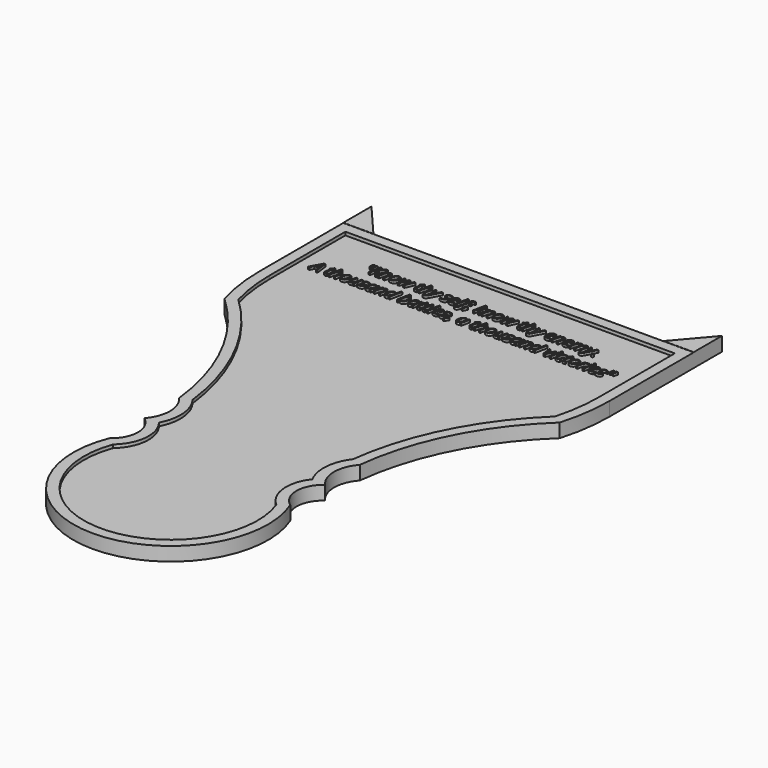
from build123d import *

# Parameters (mm, degrees)
F1_DEPTH = 5
F2_T     = -3.81
F3_T     = -2.54
F6_DEPTH = 5.08
F7_DEPTH = 5.08
F9_DEPTH = 0.8636


# Not quite as in the source:
# - the program builds the solid bodies; features that only make, move or delete a surface that nothing else refers to are left out


with BuildPart() as f1:
    # F0 (on Top) → F1 (new body)
    with BuildSketch(Plane.XY):
        with BuildLine():
            Line((52.5886416435, 57.2558040679), (0, 57.2558040679))
            Line((0, 57.2558040679), (-52.5886416435, 57.2558040679))
            Line((-52.5886416435, 57.2558040679), (-63.5, 57.2558040679))
            Line((-63.5, 57.2558040679), (-63.5, 19.1558040679))
            ThreePointArc((-63.5, 19.1558040679), (-62.8068475229, 9.4791064098), (-60.7415437698, 0))
            ThreePointArc((-60.7415437698, 0), (-41.7627075808, -25.2793542976), (-32.7543020248, -55.5793642998))
            ThreePointArc((-32.7543020248, -55.5793642998), (-29.7431167323, -63.4575262666), (-32.7543020248, -71.3356882334))
            ThreePointArc((-32.7543020248, -71.3356882334), (-28.7262743829, -79.2096882334), (-32.7543020248, -87.0836882334))
            ThreePointArc((-32.7543020248, -87.0836882334), (0, -135.5851108515), (32.7543020248, -87.0836882334))
            ThreePointArc((32.7543020248, -87.0836882334), (28.7262743829, -79.2096882334), (32.7543020248, -71.3356882334))
            ThreePointArc((32.7543020248, -71.3356882334), (29.7431167323, -63.4575262666), (32.7543020248, -55.5793642998))
            ThreePointArc((32.7543020248, -55.5793642998), (41.7627075808, -25.2793542976), (60.7415437698, 0))
            ThreePointArc((60.7415437698, 0), (62.8068475229, 9.4791064098), (63.5, 19.1558040679))
            Line((63.5, 19.1558040679), (63.5, 57.2558040679))
            Line((63.5, 57.2558040679), (52.5886416435, 57.2558040679))
        make_face()
    extrude(amount=F1_DEPTH)

    # F2
    f2_openings = [f1.faces().sort_by_distance(p)[0] for p in [
        (0, -21.294438, 5),
    ]]
    offset(amount=F2_T, openings=f2_openings)

    # F3
    f3_openings = [f1.faces().sort_by_distance(p)[0] for p in [
        (0, -21.294438, 0),
    ]]
    offset(amount=F3_T, openings=f3_openings, kind=Kind.INTERSECTION)

    # F0 (on Top) → F6 (join)
    with BuildSketch(Plane.XY):
        Polygon((63.5, 70.0215920806), (52.5886416435, 57.2558040679), (63.5, 57.2558040679), align=None)
    extrude(amount=F6_DEPTH)

    # F0 (on Top) → F7 (join)
    with BuildSketch(Plane.XY):
        Polygon((-63.5, 57.2558040679), (-52.5886416435, 57.2558040679), (-63.5, 70.0215920806), align=None)
    extrude(amount=F7_DEPTH)

    # F8 (on face) → F9 (join)
    with BuildSketch(Plane.XY.offset(3.81)):
        with BuildLine():
            add(Edge.make_bspline(
                [(0, 31.0147668691), (-0.4467864694, 30.5465102223), (-0.9321583328, 30.5465102223)],
                knots=[0.1659598064, 0.1659598064, 0.1659598064, 1, 1, 1], degree=2))
            Line((0, 31.0147668691), (0, 31.4675638708))
            add(Edge.make_bspline(
                [(-0.2063628382, 31.227178536), (-0.0949259668, 31.3345293887), (0, 31.4675638708)],
                knots=[0, 0, 0, 0.3951033283, 0.3951033283, 0.3951033283], degree=2))
            add(Edge.make_bspline(
                [(-0.7732730497, 30.9554753003), (-0.4884077195, 30.9554753003), (-0.2063628382, 31.227178536)],
                knots=[0, 0, 0, 1, 1, 1], degree=2))
            add(Edge.make_bspline(
                [(-1.1606146867, 31.1214117055), (-1.0224126949, 30.9554753003), (-0.7732730497, 30.9554753003)],
                knots=[0, 0, 0, 1, 1, 1], degree=2))
            add(Edge.make_bspline(
                [(-1.2988166786, 31.6220413699), (-1.2988166786, 31.2873481107), (-1.1606146867, 31.1214117055)],
                knots=[0, 0, 0, 1, 1, 1], degree=2))
            add(Edge.make_bspline(
                [(-1.1488628167, 32.5330463366), (-1.2988166786, 32.1015176681), (-1.2988166786, 31.6220413699)],
                knots=[0, 0, 0, 1, 1, 1], degree=2))
            add(Edge.make_bspline(
                [(-0.7361371403, 33.2174752486), (-0.9989089547, 32.964575005), (-1.1488628167, 32.5330463366)],
                knots=[0, 0, 0, 1, 1, 1], degree=2))
            add(Edge.make_bspline(
                [(-0.1678167044, 33.4703754922), (-0.4733653259, 33.4703754922), (-0.7361371403, 33.2174752486)],
                knots=[0, 0, 0, 1, 1, 1], degree=2))
            add(Edge.make_bspline(
                [(0, 33.4501662852), (-0.0781267156, 33.4703754922), (-0.1678167044, 33.4703754922)],
                knots=[0.6640855685, 0.6640855685, 0.6640855685, 1, 1, 1], degree=2))
            Line((0, 33.4501662852), (0, 33.8596596946))
            add(Edge.make_bspline(
                [(-0.2148241846, 33.8849814678), (-0.1023477377, 33.8849814678), (0, 33.8596596946)],
                knots=[0, 0, 0, 0.4168528014, 0.4168528014, 0.4168528014], degree=2))
            add(Edge.make_bspline(
                [(-1.0200623208, 33.5878941928), (-0.6529339003, 33.8849814678), (-0.2148241846, 33.8849814678)],
                knots=[0, 0, 0, 1, 1, 1], degree=2))
            add(Edge.make_bspline(
                [(-1.5959039536, 32.7680837377), (-1.3871907414, 33.2908069178), (-1.0200623208, 33.5878941928)],
                knots=[0, 0, 0, 1, 1, 1], degree=2))
            add(Edge.make_bspline(
                [(-1.8046171658, 31.6342633147), (-1.8046171658, 32.2453605576), (-1.5959039536, 32.7680837377)],
                knots=[0, 0, 0, 1, 1, 1], degree=2))
            add(Edge.make_bspline(
                [(-1.5724002135, 30.8374865249), (-1.8046171658, 31.1284628275), (-1.8046171658, 31.6342633147)],
                knots=[0, 0, 0, 1, 1, 1], degree=2))
            add(Edge.make_bspline(
                [(-0.9321583328, 30.5465102223), (-1.3401832612, 30.5465102223), (-1.5724002135, 30.8374865249)],
                knots=[0, 0, 0, 1, 1, 1], degree=2))
        make_face()
        with BuildLine():
            Line((0, 31.4675638708), (0, 31.0147668691))
            add(Edge.make_bspline(
                [(0.1762780508, 31.2196573391), (0.0889029049, 31.1079419739), (0, 31.0147668691)],
                knots=[0, 0, 0, 0.1659598064, 0.1659598064, 0.1659598064], degree=2))
            Line((0.1762780508, 31.2196573391), (0.1997817909, 31.2196573391))
            Line((0.1997817909, 31.2196573391), (0.1226895234, 30.6057396474))
            Line((0.1226895234, 30.6057396474), (0.5137917588, 30.6057396474))
            Line((0.5137917588, 30.6057396474), (1.1982206709, 33.8257520427))
            Line((1.1982206709, 33.8257520427), (0.8249812779, 33.8257520427))
            Line((0.8249812779, 33.8257520427), (0.6284900106, 33.3208917051))
            Line((0.6284900106, 33.3208917051), (0.5955847744, 33.3208917051))
            add(Edge.make_bspline(
                [(0.2665324129, 33.7392582791), (0.4780660739, 33.5935350904), (0.5955847744, 33.3208917051)],
                knots=[0, 0, 0, 1, 1, 1], degree=2))
            add(Edge.make_bspline(
                [(0, 33.8596596946), (0.143177151, 33.8242363484), (0.2665324129, 33.7392582791)],
                knots=[0.4168528014, 0.4168528014, 0.4168528014, 1, 1, 1], degree=2))
            Line((0, 33.8596596946), (0, 33.4501662852))
            add(Edge.make_bspline(
                [(0.2637119641, 33.2912769926), (0.1544525018, 33.4102137216), (0, 33.4501662852)],
                knots=[0, 0, 0, 0.6640855685, 0.6640855685, 0.6640855685], degree=2))
            add(Edge.make_bspline(
                [(0.4282381448, 32.8094503203), (0.4282381448, 33.1121784929), (0.2637119641, 33.2912769926)],
                knots=[0, 0, 0, 1, 1, 1], degree=2))
            add(Edge.make_bspline(
                [(0.251960094, 31.9351111881), (0.4282381448, 32.3713406046), (0.4282381448, 32.8094503203)],
                knots=[0, 0, 0, 1, 1, 1], degree=2))
            add(Edge.make_bspline(
                [(0, 31.4675638708), (0.1453300878, 31.671237466), (0.251960094, 31.9351111881)],
                knots=[0.3951033283, 0.3951033283, 0.3951033283, 1, 1, 1], degree=2))
        make_face()
        with BuildLine():
            Line((-0.6143877665, 40.3287668568), (0, 38.9576944297))
            Line((0, 38.9576944297), (0, 40.1223718637))
            Line((0, 40.1223718637), (-0.2411483735, 40.6371359271))
            Line((-0.2411483735, 40.6371359271), (0, 40.8772966623))
            Line((0, 40.8772966623), (0, 41.4517704126))
            Line((0, 41.4517704126), (-0.9998491044, 40.4312431637))
            Line((-0.9998491044, 40.4312431637), (-1.0111308996, 40.4312431637))
            add(Edge.make_bspline(
                [(-0.7116932506, 41.5918578505), (-0.879509955, 40.8101234543), (-1.0111308996, 40.4312431637)],
                knots=[0, 0, 0, 1, 1, 1], degree=2))
            add(Edge.make_bspline(
                [(-0.3323428852, 43.3607493313), (-0.5438765462, 42.3735922466), (-0.7116932506, 41.5918578505)],
                knots=[0, 0, 0, 1, 1, 1], degree=2))
            Line((-0.3323428852, 43.3607493313), (-0.8325024748, 43.3607493313))
            Line((-0.8325024748, 43.3607493313), (-1.801796717, 38.7888018047))
            Line((-1.801796717, 38.7888018047), (-1.302577277, 38.7888018047))
            Line((-1.302577277, 38.7888018047), (-1.0609588286, 39.9668092591))
            Line((-1.0609588286, 39.9668092591), (-0.6143877665, 40.3287668568))
        make_face()
        Polygon((0, 40.1223718637), (0, 38.9576944297), (0.0756820432, 38.7888018047), (0.6247294122, 38.7888018047), align=None)
        Polygon((-0.2411483735, 40.6371359271), (0, 40.1223718637), (0, 40.8772966623), align=None)
        Polygon((0, 41.4517704126), (0, 40.8772966623), (1.136170797, 42.0088142), (0.5457568454, 42.0088142), align=None)
        Polygon((-41.1263743727, 41.5330985002), (-40.6769828618, 43.0843453475), (-41.2297908292, 43.0843453475), (-41.4413244902, 41.5330985002), align=None)
        Polygon((-40.1044317526, 41.5330985002), (-39.6522197929, 43.0843453475), (-40.2069080595, 43.0843453475), (-40.4184417205, 41.5330985002), align=None)
        with BuildLine():
            Line((-37.2868033881, 38.7888018047), (-36.7405764679, 38.7888018047))
            Line((-36.7405764679, 38.7888018047), (-37.7681599855, 41.212507485))
            Line((-37.7681599855, 41.212507485), (-35.891621375, 43.0843453475))
            Line((-35.891621375, 43.0843453475), (-36.5055390667, 43.0843453475))
            Line((-36.5055390667, 43.0843453475), (-38.5616462517, 40.9981533752))
            Line((-38.5616462517, 40.9981533752), (-38.1178956384, 43.0843453475))
            Line((-38.1178956384, 43.0843453475), (-38.618055228, 43.0843453475))
            Line((-38.618055228, 43.0843453475), (-39.5252995963, 38.7888018047))
            Line((-39.5252995963, 38.7888018047), (-39.0260801563, 38.7888018047))
            Line((-39.0260801563, 38.7888018047), (-38.658481661, 40.5224376754))
            Line((-38.658481661, 40.5224376754), (-38.1479804257, 40.9069588636))
            add(Edge.make_bspline(
                [(-37.7173919069, 39.8450598853), (-37.9364467647, 40.3691932898), (-38.1479804257, 40.9069588636)],
                knots=[0, 0, 0, 1, 1, 1], degree=2))
            add(Edge.make_bspline(
                [(-37.2868033881, 38.7888018047), (-37.4983370491, 39.3209264809), (-37.7173919069, 39.8450598853)],
                knots=[0, 0, 0, 1, 1, 1], degree=2))
        make_face()
        with BuildLine():
            Line((-33.8486762845, 40.8223453992), (-34.2839655514, 38.7888018047))
            Line((-34.2839655514, 38.7888018047), (-33.7847461114, 38.7888018047))
            Line((-33.7847461114, 38.7888018047), (-33.3644992382, 40.7631159741))
            add(Edge.make_bspline(
                [(-33.2968084667, 41.2924202014), (-33.2968084667, 41.0602032491), (-33.3644992382, 40.7631159741)],
                knots=[0, 0, 0, 1, 1, 1], degree=2))
            add(Edge.make_bspline(
                [(-33.5125728009, 41.8635610861), (-33.2968084667, 41.6590785472), (-33.2968084667, 41.2924202014)],
                knots=[0, 0, 0, 1, 1, 1], degree=2))
            add(Edge.make_bspline(
                [(-34.1015765281, 42.0680436251), (-33.7283371351, 42.0680436251), (-33.5125728009, 41.8635610861)],
                knots=[0, 0, 0, 1, 1, 1], degree=2))
            add(Edge.make_bspline(
                [(-34.6463932239, 41.9194999876), (-34.3836214094, 42.0680436251), (-34.1015765281, 42.0680436251)],
                knots=[0, 0, 0, 1, 1, 1], degree=2))
            add(Edge.make_bspline(
                [(-35.1912099197, 41.4127593508), (-34.9091650383, 41.7709563501), (-34.6463932239, 41.9194999876)],
                knots=[0, 0, 0, 1, 1, 1], degree=2))
            Line((-35.1912099197, 41.4127593508), (-35.221294707, 41.4127593508))
            Line((-35.221294707, 41.4127593508), (-35.1564243843, 42.0088142))
            Line((-35.1564243843, 42.0088142), (-35.5644493127, 42.0088142))
            Line((-35.5644493127, 42.0088142), (-36.2526388231, 38.7888018047))
            Line((-36.2526388231, 38.7888018047), (-35.7590602808, 38.7888018047))
            Line((-35.7590602808, 38.7888018047), (-35.4619730058, 40.1839838178))
            add(Edge.make_bspline(
                [(-35.1756974512, 40.9746496351), (-35.3651375965, 40.6484177224), (-35.4619730058, 40.1839838178)],
                knots=[0, 0, 0, 1, 1, 1], degree=2))
            add(Edge.make_bspline(
                [(-34.7380578103, 41.4771595987), (-34.9862573059, 41.3008815479), (-35.1756974512, 40.9746496351)],
                knots=[0, 0, 0, 1, 1, 1], degree=2))
            add(Edge.make_bspline(
                [(-34.2275565751, 41.6534376495), (-34.4898583148, 41.6534376495), (-34.7380578103, 41.4771595987)],
                knots=[0, 0, 0, 1, 1, 1], degree=2))
            add(Edge.make_bspline(
                [(-33.8947436151, 41.5415598466), (-33.9991002212, 41.6534376495), (-34.2275565751, 41.6534376495)],
                knots=[0, 0, 0, 1, 1, 1], degree=2))
            add(Edge.make_bspline(
                [(-33.790387009, 41.2454127212), (-33.790387009, 41.4296820437), (-33.8947436151, 41.5415598466)],
                knots=[0, 0, 0, 1, 1, 1], degree=2))
            add(Edge.make_bspline(
                [(-33.8486762845, 40.8223453992), (-33.790387009, 41.1278940206), (-33.790387009, 41.2454127212)],
                knots=[0, 0, 0, 1, 1, 1], degree=2))
        make_face()
        with BuildLine():
            add(Edge.make_bspline(
                [(-31.0639531561, 42.0501807826), (-30.505504291, 42.0501807826), (-30.1820928271, 41.7197181967)],
                knots=[0, 0, 0, 1, 1, 1], degree=2))
            add(Edge.make_bspline(
                [(-31.8710715915, 41.7869388934), (-31.5067636198, 42.0501807826), (-31.0639531561, 42.0501807826)],
                knots=[0, 0, 0, 1, 1, 1], degree=2))
            add(Edge.make_bspline(
                [(-32.4502037479, 41.031998761), (-32.2353795632, 41.5236970041), (-31.8710715915, 41.7869388934)],
                knots=[0, 0, 0, 1, 1, 1], degree=2))
            add(Edge.make_bspline(
                [(-32.6650279325, 39.9818516528), (-32.6650279325, 40.5403005179), (-32.4502037479, 41.031998761)],
                knots=[0, 0, 0, 1, 1, 1], degree=2))
            add(Edge.make_bspline(
                [(-32.3444369174, 39.0736671349), (-32.6650279325, 39.4055399453), (-32.6650279325, 39.9818516528)],
                knots=[0, 0, 0, 1, 1, 1], degree=2))
            add(Edge.make_bspline(
                [(-31.4597561396, 38.7417943245), (-32.0238459022, 38.7417943245), (-32.3444369174, 39.0736671349)],
                knots=[0, 0, 0, 1, 1, 1], degree=2))
            add(Edge.make_bspline(
                [(-30.6432362081, 39.009266887), (-31.004723731, 38.7417943245), (-31.4597561396, 38.7417943245)],
                knots=[0, 0, 0, 1, 1, 1], degree=2))
            add(Edge.make_bspline(
                [(-30.0702150241, 39.767497543), (-30.2817486852, 39.2767394494), (-30.6432362081, 39.009266887)],
                knots=[0, 0, 0, 1, 1, 1], degree=2))
            add(Edge.make_bspline(
                [(-29.8586813631, 40.8101234543), (-29.8586813631, 40.2582556365), (-30.0702150241, 39.767497543)],
                knots=[0, 0, 0, 1, 1, 1], degree=2))
            add(Edge.make_bspline(
                [(-30.1820928271, 41.7197181967), (-29.8586813631, 41.3892556107), (-29.8586813631, 40.8101234543)],
                knots=[0, 0, 0, 1, 1, 1], degree=2))
        make_face()
        with BuildLine():
            add(Edge.make_bspline(
                [(-30.370122748, 40.8778142259), (-30.370122748, 41.2153279339), (-30.5539219956, 41.4254513705)],
                knots=[0, 0, 0, 1, 1, 1], degree=2))
            add(Edge.make_bspline(
                [(-30.5069145154, 39.974330456), (-30.370122748, 40.3691932898), (-30.370122748, 40.8778142259)],
                knots=[0, 0, 0, 1, 1, 1], degree=2))
            add(Edge.make_bspline(
                [(-30.8872050304, 39.3646434375), (-30.6437062829, 39.5794676221), (-30.5069145154, 39.974330456)],
                knots=[0, 0, 0, 1, 1, 1], degree=2))
            add(Edge.make_bspline(
                [(-31.4362523994, 39.1498192528), (-31.130703778, 39.1498192528), (-30.8872050304, 39.3646434375)],
                knots=[0, 0, 0, 1, 1, 1], degree=2))
            add(Edge.make_bspline(
                [(-31.9726077488, 39.3599426894), (-31.7859880523, 39.1498192528), (-31.4362523994, 39.1498192528)],
                knots=[0, 0, 0, 1, 1, 1], degree=2))
            add(Edge.make_bspline(
                [(-32.1592274453, 39.9555274639), (-32.1592274453, 39.570066126), (-31.9726077488, 39.3599426894)],
                knots=[0, 0, 0, 1, 1, 1], degree=2))
            add(Edge.make_bspline(
                [(-32.019615229, 40.8148242024), (-32.1592274453, 40.4284227149), (-32.1592274453, 39.9555274639)],
                knots=[0, 0, 0, 1, 1, 1], degree=2))
            add(Edge.make_bspline(
                [(-31.6261626195, 41.4184002484), (-31.8800030127, 41.2012256898), (-32.019615229, 40.8148242024)],
                knots=[0, 0, 0, 1, 1, 1], degree=2))
            add(Edge.make_bspline(
                [(-31.0517312112, 41.6355748071), (-31.3723222263, 41.6355748071), (-31.6261626195, 41.4184002484)],
                knots=[0, 0, 0, 1, 1, 1], degree=2))
            add(Edge.make_bspline(
                [(-30.5539219956, 41.4254513705), (-30.7377212433, 41.6355748071), (-31.0517312112, 41.6355748071)],
                knots=[0, 0, 0, 1, 1, 1], degree=2))
        make_face(mode=Mode.SUBTRACT)
        with BuildLine():
            Line((-27.2290829194, 40.5572232107), (-27.135067959, 38.7888018047))
            Line((-27.135067959, 38.7888018047), (-26.5324320625, 38.7888018047))
            Line((-26.5324320625, 38.7888018047), (-25.0460555379, 42.0088142))
            Line((-25.0460555379, 42.0088142), (-25.5687787179, 42.0088142))
            add(Edge.make_bspline(
                [(-26.5183298185, 39.8568117554), (-26.3566240865, 40.2460336917), (-25.5687787179, 42.0088142)],
                knots=[0, 0, 0, 1, 1, 1], degree=2))
            add(Edge.make_bspline(
                [(-26.761828566, 39.2146895756), (-26.6800355504, 39.4675898192), (-26.5183298185, 39.8568117554)],
                knots=[0, 0, 0, 1, 1, 1], degree=2))
            Line((-26.761828566, 39.2146895756), (-26.7796914085, 39.2146895756))
            Line((-26.7796914085, 39.2146895756), (-26.7740505109, 39.3378491737))
            Line((-26.7740505109, 39.3378491737), (-26.7740505109, 39.4939140081))
            add(Edge.make_bspline(
                [(-26.7909732038, 40.2638965341), (-26.7740505109, 39.7703179918), (-26.7740505109, 39.4939140081)],
                knots=[0, 0, 0, 1, 1, 1], degree=2))
            Line((-26.7909732038, 40.2638965341), (-26.9000305579, 42.0088142))
            Line((-26.9000305579, 42.0088142), (-27.4349756828, 42.0088142))
            Line((-27.4349756828, 42.0088142), (-28.3017936181, 40.1604800776))
            add(Edge.make_bspline(
                [(-28.7041776489, 39.2146895756), (-28.565975657, 39.5794676221), (-28.3017936181, 40.1604800776)],
                knots=[0, 0, 0, 1, 1, 1], degree=2))
            Line((-28.7041776489, 39.2146895756), (-28.7220404913, 39.2146895756))
            add(Edge.make_bspline(
                [(-28.6985367512, 40.0053553929), (-28.6985367512, 39.5728865749), (-28.7220404913, 39.2146895756)],
                knots=[0, 0, 0, 1, 1, 1], degree=2))
            Line((-28.6985367512, 40.0053553929), (-28.6985367512, 40.2638965341))
            Line((-28.6985367512, 40.2638965341), (-28.7511851291, 42.0088142))
            Line((-28.7511851291, 42.0088142), (-29.2325417266, 42.0088142))
            Line((-29.2325417266, 42.0088142), (-29.1065616796, 38.7888018047))
            Line((-29.1065616796, 38.7888018047), (-28.5133272791, 38.7888018047))
            Line((-28.5133272791, 38.7888018047), (-27.6577911391, 40.6192730846))
            Line((-27.6577911391, 40.6192730846), (-27.4142923915, 41.1749015009))
            Line((-27.4142923915, 41.1749015009), (-27.2676290532, 41.5208765553))
            Line((-27.2676290532, 41.5208765553), (-27.2413048643, 41.5208765553))
            Line((-27.2413048643, 41.5208765553), (-27.2413048643, 41.0630236979))
            add(Edge.make_bspline(
                [(-27.2290829194, 40.5572232107), (-27.2413048643, 40.8336271944), (-27.2413048643, 41.0630236979)],
                knots=[0, 0, 0, 1, 1, 1], degree=2))
        make_face()
        with BuildLine():
            add(Edge.make_bspline(
                [(-22.5396166923, 39.13289656), (-22.3779109604, 39.13289656), (-22.1165493703, 39.2090486779)],
                knots=[0, 0, 0, 1, 1, 1], degree=2))
            add(Edge.make_bspline(
                [(-22.7770044675, 39.220800548), (-22.6919209283, 39.13289656), (-22.5396166923, 39.13289656)],
                knots=[0, 0, 0, 1, 1, 1], degree=2))
            add(Edge.make_bspline(
                [(-22.8620880067, 39.4732307168), (-22.8620880067, 39.308704536), (-22.7770044675, 39.220800548)],
                knots=[0, 0, 0, 1, 1, 1], degree=2))
            add(Edge.make_bspline(
                [(-22.8094396288, 39.8615125034), (-22.8620880067, 39.605791811), (-22.8620880067, 39.4732307168)],
                knots=[0, 0, 0, 1, 1, 1], degree=2))
            Line((-22.8094396288, 39.8615125034), (-22.4305593382, 41.6355748071))
            Line((-22.4305593382, 41.6355748071), (-21.6286117256, 41.6355748071))
            Line((-21.6286117256, 41.6355748071), (-21.5524596077, 42.0088142))
            Line((-21.5524596077, 42.0088142), (-22.3572276691, 42.0088142))
            Line((-22.3572276691, 42.0088142), (-22.1955219371, 42.7496520884))
            Line((-22.1955219371, 42.7496520884), (-22.4832077161, 42.7496520884))
            Line((-22.4832077161, 42.7496520884), (-22.8508062114, 42.0793254204))
            Line((-22.8508062114, 42.0793254204), (-23.3942126828, 41.8499289169))
            Line((-23.3942126828, 41.8499289169), (-23.4355792654, 41.6355748071))
            Line((-23.4355792654, 41.6355748071), (-22.9297787782, 41.6355748071))
            Line((-22.9297787782, 41.6355748071), (-23.3030181712, 39.8671534011))
            add(Edge.make_bspline(
                [(-23.355666549, 39.4262232366), (-23.355666549, 39.6198940551), (-23.3030181712, 39.8671534011)],
                knots=[0, 0, 0, 1, 1, 1], degree=2))
            add(Edge.make_bspline(
                [(-23.1605855061, 38.9044402061), (-23.355666549, 39.0793080325), (-23.355666549, 39.4262232366)],
                knots=[0, 0, 0, 1, 1, 1], degree=2))
            add(Edge.make_bspline(
                [(-22.5979059678, 38.7295723796), (-22.9655044632, 38.7295723796), (-23.1605855061, 38.9044402061)],
                knots=[0, 0, 0, 1, 1, 1], degree=2))
            add(Edge.make_bspline(
                [(-22.3628685667, 38.7591870922), (-22.509531905, 38.7295723796), (-22.5979059678, 38.7295723796)],
                knots=[0, 0, 0, 1, 1, 1], degree=2))
            add(Edge.make_bspline(
                [(-22.1165493703, 38.8301683873), (-22.2162052284, 38.7888018047), (-22.3628685667, 38.7591870922)],
                knots=[0, 0, 0, 1, 1, 1], degree=2))
            Line((-22.1165493703, 38.8301683873), (-22.1165493703, 39.2090486779))
        make_face()
        with BuildLine():
            Line((-19.1720008091, 40.8223453992), (-19.607290076, 38.7888018047))
            Line((-19.607290076, 38.7888018047), (-19.1137115337, 38.7888018047))
            add(Edge.make_bspline(
                [(-18.6878237628, 40.7631159741), (-18.8025220146, 40.1962057626), (-19.1137115337, 38.7888018047)],
                knots=[0, 0, 0, 1, 1, 1], degree=2))
            add(Edge.make_bspline(
                [(-18.6201329913, 41.2510536188), (-18.6201329913, 41.0686645956), (-18.6878237628, 40.7631159741)],
                knots=[0, 0, 0, 1, 1, 1], degree=2))
            add(Edge.make_bspline(
                [(-18.8302564279, 41.8499289169), (-18.6201329913, 41.6383952559), (-18.6201329913, 41.2510536188)],
                knots=[0, 0, 0, 1, 1, 1], degree=2))
            add(Edge.make_bspline(
                [(-19.4249010527, 42.0614625779), (-19.0403798645, 42.0614625779), (-18.8302564279, 41.8499289169)],
                knots=[0, 0, 0, 1, 1, 1], degree=2))
            add(Edge.make_bspline(
                [(-19.987580591, 41.9058678183), (-19.7191678789, 42.0614625779), (-19.4249010527, 42.0614625779)],
                knots=[0, 0, 0, 1, 1, 1], degree=2))
            add(Edge.make_bspline(
                [(-20.5323972868, 41.3892556107), (-20.2559933031, 41.7502730588), (-19.987580591, 41.9058678183)],
                knots=[0, 0, 0, 1, 1, 1], degree=2))
            Line((-20.5323972868, 41.3892556107), (-20.565302523, 41.3892556107))
            add(Edge.make_bspline(
                [(-20.4252202319, 41.9439438773), (-20.4853898066, 41.6882231849), (-20.565302523, 41.3892556107)],
                knots=[0, 0, 0, 1, 1, 1], degree=2))
            add(Edge.make_bspline(
                [(-20.3138125038, 42.4332917465), (-20.3650506572, 42.1996645697), (-20.4252202319, 41.9439438773)],
                knots=[0, 0, 0, 1, 1, 1], degree=2))
            add(Edge.make_bspline(
                [(-20.2141566457, 42.893024903), (-20.2625743503, 42.6669189232), (-20.3138125038, 42.4332917465)],
                knots=[0, 0, 0, 1, 1, 1], degree=2))
            add(Edge.make_bspline(
                [(-20.1121504136, 43.3607493313), (-20.1657389411, 43.1191308829), (-20.2141566457, 42.893024903)],
                knots=[0, 0, 0, 1, 1, 1], degree=2))
            Line((-20.1121504136, 43.3607493313), (-20.605728956, 43.3607493313))
            Line((-20.605728956, 43.3607493313), (-21.5759633478, 38.7888018047))
            Line((-21.5759633478, 38.7888018047), (-21.0823848054, 38.7888018047))
            Line((-21.0823848054, 38.7888018047), (-20.7852975304, 40.1783429201))
            add(Edge.make_bspline(
                [(-20.4990219758, 40.9760598595), (-20.6884621211, 40.6455972736), (-20.7852975304, 40.1783429201)],
                knots=[0, 0, 0, 1, 1, 1], degree=2))
            add(Edge.make_bspline(
                [(-20.061382335, 41.4799800475), (-20.3095818305, 41.3065224455), (-20.4990219758, 40.9760598595)],
                knots=[0, 0, 0, 1, 1, 1], degree=2))
            add(Edge.make_bspline(
                [(-19.5508810997, 41.6534376495), (-19.8131828394, 41.6534376495), (-20.061382335, 41.4799800475)],
                knots=[0, 0, 0, 1, 1, 1], degree=2))
            add(Edge.make_bspline(
                [(-19.1193524313, 41.2181483827), (-19.1193524313, 41.6534376495), (-19.5508810997, 41.6534376495)],
                knots=[0, 0, 0, 1, 1, 1], degree=2))
            add(Edge.make_bspline(
                [(-19.1720008091, 40.8223453992), (-19.1193524313, 41.0978092333), (-19.1193524313, 41.2181483827)],
                knots=[0, 0, 0, 1, 1, 1], degree=2))
        make_face()
        with BuildLine():
            Line((-17.4947739148, 42.0088142), (-17.9883524571, 42.0088142))
            Line((-17.9883524571, 42.0088142), (-17.5004148124, 38.7361534269))
            Line((-17.5004148124, 38.7361534269), (-17.7232302687, 38.336589845))
            add(Edge.make_bspline(
                [(-18.0569833782, 37.8970699049), (-17.8849360006, 38.0451434676), (-17.7232302687, 38.336589845)],
                knots=[0, 0, 0, 1, 1, 1], degree=2))
            add(Edge.make_bspline(
                [(-18.4697090546, 37.7489963422), (-18.2290307559, 37.7489963422), (-18.0569833782, 37.8970699049)],
                knots=[0, 0, 0, 1, 1, 1], degree=2))
            add(Edge.make_bspline(
                [(-18.8551703924, 37.80164472), (-18.6699609204, 37.7489963422), (-18.4697090546, 37.7489963422)],
                knots=[0, 0, 0, 1, 1, 1], degree=2))
            Line((-18.8551703924, 37.80164472), (-18.8551703924, 37.4049015869))
            add(Edge.make_bspline(
                [(-18.4433848657, 37.3428517131), (-18.6549185267, 37.3428517131), (-18.8551703924, 37.4049015869)],
                knots=[0, 0, 0, 1, 1, 1], degree=2))
            add(Edge.make_bspline(
                [(-17.7998524614, 37.5398130552), (-18.0673250239, 37.3428517131), (-18.4433848657, 37.3428517131)],
                knots=[0, 0, 0, 1, 1, 1], degree=2))
            add(Edge.make_bspline(
                [(-17.2597365136, 38.2425748845), (-17.5323798989, 37.7367743973), (-17.7998524614, 37.5398130552)],
                knots=[0, 0, 0, 1, 1, 1], degree=2))
            Line((-17.2597365136, 38.2425748845), (-15.2149111239, 42.0088142))
            Line((-15.2149111239, 42.0088142), (-15.737634304, 42.0088142))
            Line((-15.737634304, 42.0088142), (-16.6928263022, 40.2197095027))
            add(Edge.make_bspline(
                [(-16.918932282, 39.7613865706), (-16.7661579713, 40.0937294557), (-16.6928263022, 40.2197095027)],
                knots=[0, 0, 0, 1, 1, 1], degree=2))
            add(Edge.make_bspline(
                [(-17.1741828996, 39.173322993), (-17.0717065928, 39.4290436854), (-16.918932282, 39.7613865706)],
                knots=[0, 0, 0, 1, 1, 1], degree=2))
            Line((-17.1741828996, 39.173322993), (-17.1920457421, 39.173322993))
            add(Edge.make_bspline(
                [(-17.2197801555, 39.8098042752), (-17.1920457421, 39.4149414413), (-17.1920457421, 39.173322993)],
                knots=[0, 0, 0, 1, 1, 1], degree=2))
            add(Edge.make_bspline(
                [(-17.2766592065, 40.4077394236), (-17.2475145688, 40.2046671091), (-17.2197801555, 39.8098042752)],
                knots=[0, 0, 0, 1, 1, 1], degree=2))
            Line((-17.2766592065, 40.4077394236), (-17.4947739148, 42.0088142))
        make_face()
        with BuildLine():
            add(Edge.make_bspline(
                [(-11.7739635716, 39.7026272203), (-11.7739635716, 39.2438342133), (-12.0987852599, 38.9867032965)],
                knots=[0, 0, 0, 1, 1, 1], degree=2))
            add(Edge.make_bspline(
                [(-11.8416543431, 40.0302693574), (-11.7739635716, 39.8850162435), (-11.7739635716, 39.7026272203)],
                knots=[0, 0, 0, 1, 1, 1], degree=2))
            add(Edge.make_bspline(
                [(-12.0456668073, 40.3019725931), (-11.9093451146, 40.1755224713), (-11.8416543431, 40.0302693574)],
                knots=[0, 0, 0, 1, 1, 1], degree=2))
            add(Edge.make_bspline(
                [(-12.4969386174, 40.604230691), (-12.1819884999, 40.4284227149), (-12.0456668073, 40.3019725931)],
                knots=[0, 0, 0, 1, 1, 1], degree=2))
            add(Edge.make_bspline(
                [(-12.9275271363, 40.9069588636), (-12.8231705302, 40.789440163), (-12.4969386174, 40.604230691)],
                knots=[0, 0, 0, 1, 1, 1], degree=2))
            add(Edge.make_bspline(
                [(-13.0318837423, 41.1890037449), (-13.0318837423, 41.0244775642), (-12.9275271363, 40.9069588636)],
                knots=[0, 0, 0, 1, 1, 1], degree=2))
            add(Edge.make_bspline(
                [(-12.875818908, 41.5199364057), (-13.0318837423, 41.3920760595), (-13.0318837423, 41.1890037449)],
                knots=[0, 0, 0, 1, 1, 1], degree=2))
            add(Edge.make_bspline(
                [(-12.4471106884, 41.6477967519), (-12.7197540737, 41.6477967519), (-12.875818908, 41.5199364057)],
                knots=[0, 0, 0, 1, 1, 1], degree=2))
            add(Edge.make_bspline(
                [(-11.8002877605, 41.5208765553), (-12.0973750355, 41.6477967519), (-12.4471106884, 41.6477967519)],
                knots=[0, 0, 0, 1, 1, 1], degree=2))
            Line((-11.8002877605, 41.5208765553), (-11.6357615797, 41.4475448862))
            Line((-11.6357615797, 41.4475448862), (-11.4768762966, 41.8499289169))
            add(Edge.make_bspline(
                [(-12.4471106884, 42.0680436251), (-11.94413065, 42.0680436251), (-11.4768762966, 41.8499289169)],
                knots=[0, 0, 0, 1, 1, 1], degree=2))
            add(Edge.make_bspline(
                [(-13.2283750097, 41.8193740547), (-12.9312877347, 42.0680436251), (-12.4471106884, 42.0680436251)],
                knots=[0, 0, 0, 1, 1, 1], degree=2))
            add(Edge.make_bspline(
                [(-13.5254622847, 41.1655000048), (-13.5254622847, 41.5707044844), (-13.2283750097, 41.8193740547)],
                knots=[0, 0, 0, 1, 1, 1], degree=2))
            add(Edge.make_bspline(
                [(-13.3665770015, 40.6780324349), (-13.5254622847, 40.8834551235), (-13.5254622847, 41.1655000048)],
                knots=[0, 0, 0, 1, 1, 1], degree=2))
            add(Edge.make_bspline(
                [(-12.825990979, 40.2582556365), (-13.2076917184, 40.4726097463), (-13.3665770015, 40.6780324349)],
                knots=[0, 0, 0, 1, 1, 1], degree=2))
            add(Edge.make_bspline(
                [(-12.3822403657, 39.943305519), (-12.4847166725, 40.0580037708), (-12.825990979, 40.2582556365)],
                knots=[0, 0, 0, 1, 1, 1], degree=2))
            add(Edge.make_bspline(
                [(-12.2797640588, 39.6612606377), (-12.2797640588, 39.8286072673), (-12.3822403657, 39.943305519)],
                knots=[0, 0, 0, 1, 1, 1], degree=2))
            add(Edge.make_bspline(
                [(-12.4677939797, 39.2852007959), (-12.2797640588, 39.4318641342), (-12.2797640588, 39.6612606377)],
                knots=[0, 0, 0, 1, 1, 1], degree=2))
            add(Edge.make_bspline(
                [(-13.0253026951, 39.1385374576), (-12.6558239006, 39.1385374576), (-12.4677939797, 39.2852007959)],
                knots=[0, 0, 0, 1, 1, 1], degree=2))
            add(Edge.make_bspline(
                [(-13.4662328596, 39.2062282291), (-13.2283750097, 39.1385374576), (-13.0253026951, 39.1385374576)],
                knots=[0, 0, 0, 1, 1, 1], degree=2))
            add(Edge.make_bspline(
                [(-13.9099834729, 39.3970785988), (-13.7040907095, 39.2739190006), (-13.4662328596, 39.2062282291)],
                knots=[0, 0, 0, 1, 1, 1], degree=2))
            Line((-13.9099834729, 39.3970785988), (-13.9099834729, 38.9326446942))
            add(Edge.make_bspline(
                [(-13.0140208999, 38.7295723796), (-13.510419891, 38.7295723796), (-13.9099834729, 38.9326446942)],
                knots=[0, 0, 0, 1, 1, 1], degree=2))
            add(Edge.make_bspline(
                [(-12.0987852599, 38.9867032965), (-12.4236069483, 38.7295723796), (-13.0140208999, 38.7295723796)],
                knots=[0, 0, 0, 1, 1, 1], degree=2))
        make_face()
        with BuildLine():
            add(Edge.make_bspline(
                [(-9.9105870555, 38.7295723796), (-10.4511730781, 38.7295723796), (-10.7600122232, 39.0501633948)],
                knots=[0, 0, 0, 1, 1, 1], degree=2))
            add(Edge.make_bspline(
                [(-9.4442728517, 38.7812806079), (-9.6558065127, 38.7295723796), (-9.9105870555, 38.7295723796)],
                knots=[0, 0, 0, 1, 1, 1], degree=2))
            add(Edge.make_bspline(
                [(-8.956335207, 38.961789332), (-9.2327391907, 38.8329888361), (-9.4442728517, 38.7812806079)],
                knots=[0, 0, 0, 1, 1, 1], degree=2))
            Line((-8.956335207, 38.961789332), (-8.956335207, 39.3914377012))
            add(Edge.make_bspline(
                [(-9.4423925525, 39.1972968079), (-9.2468414348, 39.2504152605), (-8.956335207, 39.3914377012)],
                knots=[0, 0, 0, 1, 1, 1], degree=2))
            add(Edge.make_bspline(
                [(-9.8231531423, 39.1441783552), (-9.6379436702, 39.1441783552), (-9.4423925525, 39.1972968079)],
                knots=[0, 0, 0, 1, 1, 1], degree=2))
            add(Edge.make_bspline(
                [(-10.382542157, 39.3604127642), (-10.2020334329, 39.1441783552), (-9.8231531423, 39.1441783552)],
                knots=[0, 0, 0, 1, 1, 1], degree=2))
            add(Edge.make_bspline(
                [(-10.563050881, 39.9611683615), (-10.563050881, 39.5766471733), (-10.382542157, 39.3604127642)],
                knots=[0, 0, 0, 1, 1, 1], degree=2))
            Line((-10.563050881, 39.9611683615), (-10.5517690858, 40.1962057626))
            Line((-10.5517690858, 40.1962057626), (-10.4549336765, 40.1962057626))
            add(Edge.make_bspline(
                [(-9.0588115139, 40.4975237109), (-9.5467491586, 40.1962057626), (-10.4549336765, 40.1962057626)],
                knots=[0, 0, 0, 1, 1, 1], degree=2))
            add(Edge.make_bspline(
                [(-8.5708738691, 41.3272057368), (-8.5708738691, 40.7988416591), (-9.0588115139, 40.4975237109)],
                knots=[0, 0, 0, 1, 1, 1], degree=2))
            add(Edge.make_bspline(
                [(-8.7974499238, 41.8724925074), (-8.5708738691, 41.6769413897), (-8.5708738691, 41.3272057368)],
                knots=[0, 0, 0, 1, 1, 1], degree=2))
            add(Edge.make_bspline(
                [(-9.4734174894, 42.0680436251), (-9.0240259785, 42.0680436251), (-8.7974499238, 41.8724925074)],
                knots=[0, 0, 0, 1, 1, 1], degree=2))
            add(Edge.make_bspline(
                [(-10.2692541296, 41.7859987438), (-9.9077666067, 42.0680436251), (-9.4734174894, 42.0680436251)],
                knots=[0, 0, 0, 1, 1, 1], degree=2))
            add(Edge.make_bspline(
                [(-10.8497965104, 40.9967431508), (-10.6307416525, 41.5039538624), (-10.2692541296, 41.7859987438)],
                knots=[0, 0, 0, 1, 1, 1], degree=2))
            add(Edge.make_bspline(
                [(-11.0688513682, 39.9376646214), (-11.0688513682, 40.4895324392), (-10.8497965104, 40.9967431508)],
                knots=[0, 0, 0, 1, 1, 1], degree=2))
            add(Edge.make_bspline(
                [(-10.7600122232, 39.0501633948), (-11.0688513682, 39.3707544099), (-11.0688513682, 39.9376646214)],
                knots=[0, 0, 0, 1, 1, 1], degree=2))
        make_face()
        with BuildLine():
            add(Edge.make_bspline(
                [(-9.5025621272, 41.6477967519), (-9.8052902998, 41.6477967519), (-10.0713526379, 41.3713927682)],
                knots=[0, 0, 0, 1, 1, 1], degree=2))
            add(Edge.make_bspline(
                [(-9.1659885688, 41.5448503702), (-9.2731656237, 41.6477967519), (-9.5025621272, 41.6477967519)],
                knots=[0, 0, 0, 1, 1, 1], degree=2))
            add(Edge.make_bspline(
                [(-9.0588115139, 41.2858391542), (-9.0588115139, 41.4419039885), (-9.1659885688, 41.5448503702)],
                knots=[0, 0, 0, 1, 1, 1], degree=2))
            add(Edge.make_bspline(
                [(-9.4160683636, 40.7790985174), (-9.0588115139, 40.9539663438), (-9.0588115139, 41.2858391542)],
                knots=[0, 0, 0, 1, 1, 1], degree=2))
            add(Edge.make_bspline(
                [(-10.4427117316, 40.604230691), (-9.7733252133, 40.604230691), (-9.4160683636, 40.7790985174)],
                knots=[0, 0, 0, 1, 1, 1], degree=2))
            Line((-10.4427117316, 40.604230691), (-10.4784374166, 40.604230691))
            add(Edge.make_bspline(
                [(-10.0713526379, 41.3713927682), (-10.3374149759, 41.0949887845), (-10.4784374166, 40.604230691)],
                knots=[0, 0, 0, 1, 1, 1], degree=2))
        make_face(mode=Mode.SUBTRACT)
        Polygon((-8.2220783659, 38.7888018047), (-7.7284998235, 38.7888018047), (-6.7526245341, 43.3607493313), (-7.2462030764, 43.3607493313), align=None)
        with BuildLine():
            add(Edge.make_bspline(
                [(-7.1672305097, 37.3428517131), (-7.3703028242, 37.3428517131), (-7.534829005, 37.4049015869)],
                knots=[0, 0, 0, 1, 1, 1], degree=2))
            add(Edge.make_bspline(
                [(-6.5410908731, 37.5985724055), (-6.778948723, 37.3428517131), (-7.1672305097, 37.3428517131)],
                knots=[0, 0, 0, 1, 1, 1], degree=2))
            add(Edge.make_bspline(
                [(-6.1885347714, 38.4099215141), (-6.3032330232, 37.8542930979), (-6.5410908731, 37.5985724055)],
                knots=[0, 0, 0, 1, 1, 1], degree=2))
            Line((-6.1885347714, 38.4099215141), (-5.5069263082, 41.6355748071))
            Line((-5.5069263082, 41.6355748071), (-4.8112156009, 41.6355748071))
            Line((-4.8112156009, 41.6355748071), (-4.7378839317, 42.0088142))
            Line((-4.7378839317, 42.0088142), (-5.4364150878, 42.0088142))
            Line((-5.4364150878, 42.0088142), (-5.3630834187, 42.3265847663))
            add(Edge.make_bspline(
                [(-5.1416781868, 42.847897722), (-5.2784699543, 42.7054650569), (-5.3630834187, 42.3265847663)],
                knots=[0, 0, 0, 1, 1, 1], degree=2))
            add(Edge.make_bspline(
                [(-4.749165727, 42.9903303871), (-5.0048864194, 42.9903303871), (-5.1416781868, 42.847897722)],
                knots=[0, 0, 0, 1, 1, 1], degree=2))
            add(Edge.make_bspline(
                [(-4.3467816963, 42.9047767731), (-4.5695971525, 42.9903303871), (-4.749165727, 42.9903303871)],
                knots=[0, 0, 0, 1, 1, 1], degree=2))
            Line((-4.3467816963, 42.9047767731), (-4.2208016493, 43.2836570637))
            add(Edge.make_bspline(
                [(-4.4849836881, 43.3588690321), (-4.3148166097, 43.3250236463), (-4.2208016493, 43.2836570637)],
                knots=[0, 0, 0, 1, 1, 1], degree=2))
            add(Edge.make_bspline(
                [(-4.7726694671, 43.3927144178), (-4.6551507665, 43.3927144178), (-4.4849836881, 43.3588690321)],
                knots=[0, 0, 0, 1, 1, 1], degree=2))
            add(Edge.make_bspline(
                [(-5.4820123437, 43.1501558199), (-5.2427442693, 43.3927144178), (-4.7726694671, 43.3927144178)],
                knots=[0, 0, 0, 1, 1, 1], degree=2))
            add(Edge.make_bspline(
                [(-5.856661961, 42.3200037191), (-5.721280418, 42.9075972219), (-5.4820123437, 43.1501558199)],
                knots=[0, 0, 0, 1, 1, 1], degree=2))
            Line((-5.856661961, 42.3200037191), (-5.9243527326, 42.0266770425))
            Line((-5.9243527326, 42.0266770425), (-6.5298090778, 41.833006224))
            Line((-6.5298090778, 41.833006224), (-6.567415062, 41.6355748071))
            Line((-6.567415062, 41.6355748071), (-6.0005048505, 41.6355748071))
            Line((-6.0005048505, 41.6355748071), (-6.6680110697, 38.4569289944))
            add(Edge.make_bspline(
                [(-6.8616818882, 37.9365561883), (-6.7413427388, 38.1184751367), (-6.6680110697, 38.4569289944)],
                knots=[0, 0, 0, 1, 1, 1], degree=2))
            add(Edge.make_bspline(
                [(-7.2057766435, 37.7546372398), (-6.9820210376, 37.7546372398), (-6.8616818882, 37.9365561883)],
                knots=[0, 0, 0, 1, 1, 1], degree=2))
            add(Edge.make_bspline(
                [(-7.534829005, 37.8195075625), (-7.3467990841, 37.7546372398), (-7.2057766435, 37.7546372398)],
                knots=[0, 0, 0, 1, 1, 1], degree=2))
            Line((-7.534829005, 37.8195075625), (-7.534829005, 37.4049015869))
        make_face()
        with BuildLine():
            Line((-4.1004624999, 39.4205823389), (-4.12396624, 39.4882731105))
            Line((-4.12396624, 39.4882731105), (-4.673013609, 39.4882731105))
            add(Edge.make_bspline(
                [(-5.2728290567, 38.013178381), (-4.9024101125, 38.8536721274), (-4.673013609, 39.4882731105)],
                knots=[0, 0, 0, 1, 1, 1], degree=2))
            Line((-5.2728290567, 38.013178381), (-4.8930086165, 38.013178381))
            add(Edge.make_bspline(
                [(-4.1004624999, 39.4205823389), (-4.4323353103, 38.7295723796), (-4.8930086165, 38.013178381)],
                knots=[0, 0, 0, 1, 1, 1], degree=2))
        make_face()
        with BuildLine():
            Line((3.5429537844, 40.8223453992), (3.1076645176, 38.7888018047))
            Line((3.1076645176, 38.7888018047), (3.6068839575, 38.7888018047))
            Line((3.6068839575, 38.7888018047), (4.0271308307, 40.7631159741))
            add(Edge.make_bspline(
                [(4.0948216023, 41.2924202014), (4.0948216023, 41.0602032491), (4.0271308307, 40.7631159741)],
                knots=[0, 0, 0, 1, 1, 1], degree=2))
            add(Edge.make_bspline(
                [(3.879057268, 41.8635610861), (4.0948216023, 41.6590785472), (4.0948216023, 41.2924202014)],
                knots=[0, 0, 0, 1, 1, 1], degree=2))
            add(Edge.make_bspline(
                [(3.2900535408, 42.0680436251), (3.6632929338, 42.0680436251), (3.879057268, 41.8635610861)],
                knots=[0, 0, 0, 1, 1, 1], degree=2))
            add(Edge.make_bspline(
                [(2.745236845, 41.9194999876), (3.0080086595, 42.0680436251), (3.2900535408, 42.0680436251)],
                knots=[0, 0, 0, 1, 1, 1], degree=2))
            add(Edge.make_bspline(
                [(2.2004201493, 41.4127593508), (2.4824650306, 41.7709563501), (2.745236845, 41.9194999876)],
                knots=[0, 0, 0, 1, 1, 1], degree=2))
            Line((2.2004201493, 41.4127593508), (2.1703353619, 41.4127593508))
            Line((2.1703353619, 41.4127593508), (2.2352056846, 42.0088142))
            Line((2.2352056846, 42.0088142), (1.8271807563, 42.0088142))
            Line((1.8271807563, 42.0088142), (1.1389912458, 38.7888018047))
            Line((1.1389912458, 38.7888018047), (1.6325697882, 38.7888018047))
            Line((1.6325697882, 38.7888018047), (1.9296570632, 40.1839838178))
            add(Edge.make_bspline(
                [(2.2159326177, 40.9746496351), (2.0264924724, 40.6484177224), (1.9296570632, 40.1839838178)],
                knots=[0, 0, 0, 1, 1, 1], degree=2))
            add(Edge.make_bspline(
                [(2.6535722586, 41.4771595987), (2.405372763, 41.3008815479), (2.2159326177, 40.9746496351)],
                knots=[0, 0, 0, 1, 1, 1], degree=2))
            add(Edge.make_bspline(
                [(3.1640734938, 41.6534376495), (2.9017717542, 41.6534376495), (2.6535722586, 41.4771595987)],
                knots=[0, 0, 0, 1, 1, 1], degree=2))
            add(Edge.make_bspline(
                [(3.4968864538, 41.5415598466), (3.3925298477, 41.6534376495), (3.1640734938, 41.6534376495)],
                knots=[0, 0, 0, 1, 1, 1], degree=2))
            add(Edge.make_bspline(
                [(3.6012430599, 41.2454127212), (3.6012430599, 41.4296820437), (3.4968864538, 41.5415598466)],
                knots=[0, 0, 0, 1, 1, 1], degree=2))
            add(Edge.make_bspline(
                [(3.5429537844, 40.8223453992), (3.6012430599, 41.1278940206), (3.6012430599, 41.2454127212)],
                knots=[0, 0, 0, 1, 1, 1], degree=2))
        make_face()
        with BuildLine():
            add(Edge.make_bspline(
                [(6.3276769129, 42.0501807826), (6.8861257779, 42.0501807826), (7.2095372419, 41.7197181967)],
                knots=[0, 0, 0, 1, 1, 1], degree=2))
            add(Edge.make_bspline(
                [(5.5205584774, 41.7869388934), (5.8848664492, 42.0501807826), (6.3276769129, 42.0501807826)],
                knots=[0, 0, 0, 1, 1, 1], degree=2))
            add(Edge.make_bspline(
                [(4.9414263211, 41.031998761), (5.1562505057, 41.5236970041), (5.5205584774, 41.7869388934)],
                knots=[0, 0, 0, 1, 1, 1], degree=2))
            add(Edge.make_bspline(
                [(4.7266021365, 39.9818516528), (4.7266021365, 40.5403005179), (4.9414263211, 41.031998761)],
                knots=[0, 0, 0, 1, 1, 1], degree=2))
            add(Edge.make_bspline(
                [(5.0471931516, 39.0736671349), (4.7266021365, 39.4055399453), (4.7266021365, 39.9818516528)],
                knots=[0, 0, 0, 1, 1, 1], degree=2))
            add(Edge.make_bspline(
                [(5.9318739294, 38.7417943245), (5.3677841667, 38.7417943245), (5.0471931516, 39.0736671349)],
                knots=[0, 0, 0, 1, 1, 1], degree=2))
            add(Edge.make_bspline(
                [(6.7483938609, 39.009266887), (6.386906338, 38.7417943245), (5.9318739294, 38.7417943245)],
                knots=[0, 0, 0, 1, 1, 1], degree=2))
            add(Edge.make_bspline(
                [(7.3214150448, 39.767497543), (7.1098813838, 39.2767394494), (6.7483938609, 39.009266887)],
                knots=[0, 0, 0, 1, 1, 1], degree=2))
            add(Edge.make_bspline(
                [(7.5329487058, 40.8101234543), (7.5329487058, 40.2582556365), (7.3214150448, 39.767497543)],
                knots=[0, 0, 0, 1, 1, 1], degree=2))
            add(Edge.make_bspline(
                [(7.2095372419, 41.7197181967), (7.5329487058, 41.3892556107), (7.5329487058, 40.8101234543)],
                knots=[0, 0, 0, 1, 1, 1], degree=2))
        make_face()
        with BuildLine():
            add(Edge.make_bspline(
                [(7.021507321, 40.8778142259), (7.021507321, 41.2153279339), (6.8377080733, 41.4254513705)],
                knots=[0, 0, 0, 1, 1, 1], degree=2))
            add(Edge.make_bspline(
                [(6.8847155535, 39.974330456), (7.021507321, 40.3691932898), (7.021507321, 40.8778142259)],
                knots=[0, 0, 0, 1, 1, 1], degree=2))
            add(Edge.make_bspline(
                [(6.5044250385, 39.3646434375), (6.7479237861, 39.5794676221), (6.8847155535, 39.974330456)],
                knots=[0, 0, 0, 1, 1, 1], degree=2))
            add(Edge.make_bspline(
                [(5.9553776695, 39.1498192528), (6.260926291, 39.1498192528), (6.5044250385, 39.3646434375)],
                knots=[0, 0, 0, 1, 1, 1], degree=2))
            add(Edge.make_bspline(
                [(5.4190223202, 39.3599426894), (5.6056420166, 39.1498192528), (5.9553776695, 39.1498192528)],
                knots=[0, 0, 0, 1, 1, 1], degree=2))
            add(Edge.make_bspline(
                [(5.2324026237, 39.9555274639), (5.2324026237, 39.570066126), (5.4190223202, 39.3599426894)],
                knots=[0, 0, 0, 1, 1, 1], degree=2))
            add(Edge.make_bspline(
                [(5.3720148399, 40.8148242024), (5.2324026237, 40.4284227149), (5.2324026237, 39.9555274639)],
                knots=[0, 0, 0, 1, 1, 1], degree=2))
            add(Edge.make_bspline(
                [(5.7654674494, 41.4184002484), (5.5116270562, 41.2012256898), (5.3720148399, 40.8148242024)],
                knots=[0, 0, 0, 1, 1, 1], degree=2))
            add(Edge.make_bspline(
                [(6.3398988577, 41.6355748071), (6.0193078426, 41.6355748071), (5.7654674494, 41.4184002484)],
                knots=[0, 0, 0, 1, 1, 1], degree=2))
            add(Edge.make_bspline(
                [(6.8377080733, 41.4254513705), (6.6539088256, 41.6355748071), (6.3398988577, 41.6355748071)],
                knots=[0, 0, 0, 1, 1, 1], degree=2))
        make_face(mode=Mode.SUBTRACT)
        with BuildLine():
            Line((10.1625471495, 40.5572232107), (10.25656211, 38.7888018047))
            Line((10.25656211, 38.7888018047), (10.8591980064, 38.7888018047))
            Line((10.8591980064, 38.7888018047), (12.3455745311, 42.0088142))
            Line((12.3455745311, 42.0088142), (11.822851351, 42.0088142))
            add(Edge.make_bspline(
                [(10.8733002505, 39.8568117554), (11.0350059825, 40.2460336917), (11.822851351, 42.0088142)],
                knots=[0, 0, 0, 1, 1, 1], degree=2))
            add(Edge.make_bspline(
                [(10.6298015029, 39.2146895756), (10.7115945185, 39.4675898192), (10.8733002505, 39.8568117554)],
                knots=[0, 0, 0, 1, 1, 1], degree=2))
            Line((10.6298015029, 39.2146895756), (10.6119386604, 39.2146895756))
            Line((10.6119386604, 39.2146895756), (10.6175795581, 39.3378491737))
            Line((10.6175795581, 39.3378491737), (10.6175795581, 39.4939140081))
            add(Edge.make_bspline(
                [(10.6006568652, 40.2638965341), (10.6175795581, 39.7703179918), (10.6175795581, 39.4939140081)],
                knots=[0, 0, 0, 1, 1, 1], degree=2))
            Line((10.6006568652, 40.2638965341), (10.4915995111, 42.0088142))
            Line((10.4915995111, 42.0088142), (9.9566543861, 42.0088142))
            Line((9.9566543861, 42.0088142), (9.0898364508, 40.1604800776))
            add(Edge.make_bspline(
                [(8.6874524201, 39.2146895756), (8.825654412, 39.5794676221), (9.0898364508, 40.1604800776)],
                knots=[0, 0, 0, 1, 1, 1], degree=2))
            Line((8.6874524201, 39.2146895756), (8.6695895776, 39.2146895756))
            add(Edge.make_bspline(
                [(8.6930933177, 40.0053553929), (8.6930933177, 39.5728865749), (8.6695895776, 39.2146895756)],
                knots=[0, 0, 0, 1, 1, 1], degree=2))
            Line((8.6930933177, 40.0053553929), (8.6930933177, 40.2638965341))
            Line((8.6930933177, 40.2638965341), (8.6404449399, 42.0088142))
            Line((8.6404449399, 42.0088142), (8.1590883424, 42.0088142))
            Line((8.1590883424, 42.0088142), (8.2850683894, 38.7888018047))
            Line((8.2850683894, 38.7888018047), (8.8783027898, 38.7888018047))
            Line((8.8783027898, 38.7888018047), (9.7338389299, 40.6192730846))
            Line((9.7338389299, 40.6192730846), (9.9773376774, 41.1749015009))
            Line((9.9773376774, 41.1749015009), (10.1240010157, 41.5208765553))
            Line((10.1240010157, 41.5208765553), (10.1503252047, 41.5208765553))
            Line((10.1503252047, 41.5208765553), (10.1503252047, 41.0630236979))
            add(Edge.make_bspline(
                [(10.1625471495, 40.5572232107), (10.1503252047, 40.8336271944), (10.1503252047, 41.0630236979)],
                knots=[0, 0, 0, 1, 1, 1], degree=2))
        make_face()
        with BuildLine():
            add(Edge.make_bspline(
                [(14.8520133766, 39.13289656), (15.0137191086, 39.13289656), (15.2750806986, 39.2090486779)],
                knots=[0, 0, 0, 1, 1, 1], degree=2))
            add(Edge.make_bspline(
                [(14.6146256015, 39.220800548), (14.6997091407, 39.13289656), (14.8520133766, 39.13289656)],
                knots=[0, 0, 0, 1, 1, 1], degree=2))
            add(Edge.make_bspline(
                [(14.5295420623, 39.4732307168), (14.5295420623, 39.308704536), (14.6146256015, 39.220800548)],
                knots=[0, 0, 0, 1, 1, 1], degree=2))
            add(Edge.make_bspline(
                [(14.5821904401, 39.8615125034), (14.5295420623, 39.605791811), (14.5295420623, 39.4732307168)],
                knots=[0, 0, 0, 1, 1, 1], degree=2))
            Line((14.5821904401, 39.8615125034), (14.9610707307, 41.6355748071))
            Line((14.9610707307, 41.6355748071), (15.7630183433, 41.6355748071))
            Line((15.7630183433, 41.6355748071), (15.8391704613, 42.0088142))
            Line((15.8391704613, 42.0088142), (15.0344023999, 42.0088142))
            Line((15.0344023999, 42.0088142), (15.1961081318, 42.7496520884))
            Line((15.1961081318, 42.7496520884), (14.9084223529, 42.7496520884))
            Line((14.9084223529, 42.7496520884), (14.5408238575, 42.0793254204))
            Line((14.5408238575, 42.0793254204), (13.9974173861, 41.8499289169))
            Line((13.9974173861, 41.8499289169), (13.9560508035, 41.6355748071))
            Line((13.9560508035, 41.6355748071), (14.4618512907, 41.6355748071))
            Line((14.4618512907, 41.6355748071), (14.0886118978, 39.8671534011))
            add(Edge.make_bspline(
                [(14.0359635199, 39.4262232366), (14.0359635199, 39.6198940551), (14.0886118978, 39.8671534011)],
                knots=[0, 0, 0, 1, 1, 1], degree=2))
            add(Edge.make_bspline(
                [(14.2310445629, 38.9044402061), (14.0359635199, 39.0793080325), (14.0359635199, 39.4262232366)],
                knots=[0, 0, 0, 1, 1, 1], degree=2))
            add(Edge.make_bspline(
                [(14.7937241011, 38.7295723796), (14.4261256058, 38.7295723796), (14.2310445629, 38.9044402061)],
                knots=[0, 0, 0, 1, 1, 1], degree=2))
            add(Edge.make_bspline(
                [(15.0287615022, 38.7591870922), (14.8820981639, 38.7295723796), (14.7937241011, 38.7295723796)],
                knots=[0, 0, 0, 1, 1, 1], degree=2))
            add(Edge.make_bspline(
                [(15.2750806986, 38.8301683873), (15.1754248405, 38.7888018047), (15.0287615022, 38.7591870922)],
                knots=[0, 0, 0, 1, 1, 1], degree=2))
            Line((15.2750806986, 38.8301683873), (15.2750806986, 39.2090486779))
        make_face()
        with BuildLine():
            Line((18.2196292598, 40.8223453992), (17.7843399929, 38.7888018047))
            Line((17.7843399929, 38.7888018047), (18.2779185353, 38.7888018047))
            add(Edge.make_bspline(
                [(18.7038063061, 40.7631159741), (18.5891080544, 40.1962057626), (18.2779185353, 38.7888018047)],
                knots=[0, 0, 0, 1, 1, 1], degree=2))
            add(Edge.make_bspline(
                [(18.7714970776, 41.2510536188), (18.7714970776, 41.0686645956), (18.7038063061, 40.7631159741)],
                knots=[0, 0, 0, 1, 1, 1], degree=2))
            add(Edge.make_bspline(
                [(18.561373641, 41.8499289169), (18.7714970776, 41.6383952559), (18.7714970776, 41.2510536188)],
                knots=[0, 0, 0, 1, 1, 1], degree=2))
            add(Edge.make_bspline(
                [(17.9667290162, 42.0614625779), (18.3512502044, 42.0614625779), (18.561373641, 41.8499289169)],
                knots=[0, 0, 0, 1, 1, 1], degree=2))
            add(Edge.make_bspline(
                [(17.4040494779, 41.9058678183), (17.67246219, 42.0614625779), (17.9667290162, 42.0614625779)],
                knots=[0, 0, 0, 1, 1, 1], degree=2))
            add(Edge.make_bspline(
                [(16.8592327821, 41.3892556107), (17.1356367659, 41.7502730588), (17.4040494779, 41.9058678183)],
                knots=[0, 0, 0, 1, 1, 1], degree=2))
            Line((16.8592327821, 41.3892556107), (16.826327546, 41.3892556107))
            add(Edge.make_bspline(
                [(16.9664098371, 41.9439438773), (16.9062402624, 41.6882231849), (16.826327546, 41.3892556107)],
                knots=[0, 0, 0, 1, 1, 1], degree=2))
            add(Edge.make_bspline(
                [(17.0778175652, 42.4332917465), (17.0265794117, 42.1996645697), (16.9664098371, 41.9439438773)],
                knots=[0, 0, 0, 1, 1, 1], degree=2))
            add(Edge.make_bspline(
                [(17.1774734233, 42.893024903), (17.1290557186, 42.6669189232), (17.0778175652, 42.4332917465)],
                knots=[0, 0, 0, 1, 1, 1], degree=2))
            add(Edge.make_bspline(
                [(17.2794796553, 43.3607493313), (17.2258911279, 43.1191308829), (17.1774734233, 42.893024903)],
                knots=[0, 0, 0, 1, 1, 1], degree=2))
            Line((17.2794796553, 43.3607493313), (16.785901113, 43.3607493313))
            Line((16.785901113, 43.3607493313), (15.8156667212, 38.7888018047))
            Line((15.8156667212, 38.7888018047), (16.3092452635, 38.7888018047))
            Line((16.3092452635, 38.7888018047), (16.6063325385, 40.1783429201))
            add(Edge.make_bspline(
                [(16.8926080931, 40.9760598595), (16.7031679478, 40.6455972736), (16.6063325385, 40.1783429201)],
                knots=[0, 0, 0, 1, 1, 1], degree=2))
            add(Edge.make_bspline(
                [(17.330247734, 41.4799800475), (17.0820482384, 41.3065224455), (16.8926080931, 40.9760598595)],
                knots=[0, 0, 0, 1, 1, 1], degree=2))
            add(Edge.make_bspline(
                [(17.8407489692, 41.6534376495), (17.5784472296, 41.6534376495), (17.330247734, 41.4799800475)],
                knots=[0, 0, 0, 1, 1, 1], degree=2))
            add(Edge.make_bspline(
                [(18.2722776377, 41.2181483827), (18.2722776377, 41.6534376495), (17.8407489692, 41.6534376495)],
                knots=[0, 0, 0, 1, 1, 1], degree=2))
            add(Edge.make_bspline(
                [(18.2196292598, 40.8223453992), (18.2722776377, 41.0978092333), (18.2722776377, 41.2181483827)],
                knots=[0, 0, 0, 1, 1, 1], degree=2))
        make_face()
        with BuildLine():
            Line((19.8968561542, 42.0088142), (19.4032776118, 42.0088142))
            Line((19.4032776118, 42.0088142), (19.8912152566, 38.7361534269))
            Line((19.8912152566, 38.7361534269), (19.6683998003, 38.336589845))
            add(Edge.make_bspline(
                [(19.3346466907, 37.8970699049), (19.5066940683, 38.0451434676), (19.6683998003, 38.336589845)],
                knots=[0, 0, 0, 1, 1, 1], degree=2))
            add(Edge.make_bspline(
                [(18.9219210143, 37.7489963422), (19.1625993131, 37.7489963422), (19.3346466907, 37.8970699049)],
                knots=[0, 0, 0, 1, 1, 1], degree=2))
            add(Edge.make_bspline(
                [(18.5364596765, 37.80164472), (18.7216691486, 37.7489963422), (18.9219210143, 37.7489963422)],
                knots=[0, 0, 0, 1, 1, 1], degree=2))
            Line((18.5364596765, 37.80164472), (18.5364596765, 37.4049015869))
            add(Edge.make_bspline(
                [(18.9482452033, 37.3428517131), (18.7367115423, 37.3428517131), (18.5364596765, 37.4049015869)],
                knots=[0, 0, 0, 1, 1, 1], degree=2))
            add(Edge.make_bspline(
                [(19.5917776075, 37.5398130552), (19.3243050451, 37.3428517131), (18.9482452033, 37.3428517131)],
                knots=[0, 0, 0, 1, 1, 1], degree=2))
            add(Edge.make_bspline(
                [(20.1318935553, 38.2425748845), (19.85925017, 37.7367743973), (19.5917776075, 37.5398130552)],
                knots=[0, 0, 0, 1, 1, 1], degree=2))
            Line((20.1318935553, 38.2425748845), (22.176718945, 42.0088142))
            Line((22.176718945, 42.0088142), (21.6539957649, 42.0088142))
            Line((21.6539957649, 42.0088142), (20.6988037668, 40.2197095027))
            add(Edge.make_bspline(
                [(20.4726977869, 39.7613865706), (20.6254720976, 40.0937294557), (20.6988037668, 40.2197095027)],
                knots=[0, 0, 0, 1, 1, 1], degree=2))
            add(Edge.make_bspline(
                [(20.2174471693, 39.173322993), (20.3199234762, 39.4290436854), (20.4726977869, 39.7613865706)],
                knots=[0, 0, 0, 1, 1, 1], degree=2))
            Line((20.2174471693, 39.173322993), (20.1995843268, 39.173322993))
            add(Edge.make_bspline(
                [(20.1718499135, 39.8098042752), (20.1995843268, 39.4149414413), (20.1995843268, 39.173322993)],
                knots=[0, 0, 0, 1, 1, 1], degree=2))
            add(Edge.make_bspline(
                [(20.1149708624, 40.4077394236), (20.1441155002, 40.2046671091), (20.1718499135, 39.8098042752)],
                knots=[0, 0, 0, 1, 1, 1], degree=2))
            Line((20.1149708624, 40.4077394236), (19.8968561542, 42.0088142))
        make_face()
        with BuildLine():
            add(Edge.make_bspline(
                [(24.9040929476, 38.7295723796), (24.363506925, 38.7295723796), (24.0546677799, 39.0501633948)],
                knots=[0, 0, 0, 1, 1, 1], degree=2))
            add(Edge.make_bspline(
                [(25.3704071514, 38.7812806079), (25.1588734904, 38.7295723796), (24.9040929476, 38.7295723796)],
                knots=[0, 0, 0, 1, 1, 1], degree=2))
            add(Edge.make_bspline(
                [(25.8583447961, 38.961789332), (25.5819408124, 38.8329888361), (25.3704071514, 38.7812806079)],
                knots=[0, 0, 0, 1, 1, 1], degree=2))
            Line((25.8583447961, 38.961789332), (25.8583447961, 39.3914377012))
            add(Edge.make_bspline(
                [(25.3722874506, 39.1972968079), (25.5678385683, 39.2504152605), (25.8583447961, 39.3914377012)],
                knots=[0, 0, 0, 1, 1, 1], degree=2))
            add(Edge.make_bspline(
                [(24.9915268608, 39.1441783552), (25.1767363329, 39.1441783552), (25.3722874506, 39.1972968079)],
                knots=[0, 0, 0, 1, 1, 1], degree=2))
            add(Edge.make_bspline(
                [(24.4321378461, 39.3604127642), (24.6126465702, 39.1441783552), (24.9915268608, 39.1441783552)],
                knots=[0, 0, 0, 1, 1, 1], degree=2))
            add(Edge.make_bspline(
                [(24.2516291221, 39.9611683615), (24.2516291221, 39.5766471733), (24.4321378461, 39.3604127642)],
                knots=[0, 0, 0, 1, 1, 1], degree=2))
            Line((24.2516291221, 39.9611683615), (24.2629109173, 40.1962057626))
            Line((24.2629109173, 40.1962057626), (24.3597463266, 40.1962057626))
            add(Edge.make_bspline(
                [(25.7558684892, 40.4975237109), (25.2679308445, 40.1962057626), (24.3597463266, 40.1962057626)],
                knots=[0, 0, 0, 1, 1, 1], degree=2))
            add(Edge.make_bspline(
                [(26.243806134, 41.3272057368), (26.243806134, 40.7988416591), (25.7558684892, 40.4975237109)],
                knots=[0, 0, 0, 1, 1, 1], degree=2))
            add(Edge.make_bspline(
                [(26.0172300793, 41.8724925074), (26.243806134, 41.6769413897), (26.243806134, 41.3272057368)],
                knots=[0, 0, 0, 1, 1, 1], degree=2))
            add(Edge.make_bspline(
                [(25.3412625137, 42.0680436251), (25.7906540246, 42.0680436251), (26.0172300793, 41.8724925074)],
                knots=[0, 0, 0, 1, 1, 1], degree=2))
            add(Edge.make_bspline(
                [(24.5454258735, 41.7859987438), (24.9069133964, 42.0680436251), (25.3412625137, 42.0680436251)],
                knots=[0, 0, 0, 1, 1, 1], degree=2))
            add(Edge.make_bspline(
                [(23.9648834927, 40.9967431508), (24.1839383506, 41.5039538624), (24.5454258735, 41.7859987438)],
                knots=[0, 0, 0, 1, 1, 1], degree=2))
            add(Edge.make_bspline(
                [(23.7458286349, 39.9376646214), (23.7458286349, 40.4895324392), (23.9648834927, 40.9967431508)],
                knots=[0, 0, 0, 1, 1, 1], degree=2))
            add(Edge.make_bspline(
                [(24.0546677799, 39.0501633948), (23.7458286349, 39.3707544099), (23.7458286349, 39.9376646214)],
                knots=[0, 0, 0, 1, 1, 1], degree=2))
        make_face()
        with BuildLine():
            add(Edge.make_bspline(
                [(25.3121178759, 41.6477967519), (25.0093897033, 41.6477967519), (24.7433273652, 41.3713927682)],
                knots=[0, 0, 0, 1, 1, 1], degree=2))
            add(Edge.make_bspline(
                [(25.6486914343, 41.5448503702), (25.5415143794, 41.6477967519), (25.3121178759, 41.6477967519)],
                knots=[0, 0, 0, 1, 1, 1], degree=2))
            add(Edge.make_bspline(
                [(25.7558684892, 41.2858391542), (25.7558684892, 41.4419039885), (25.6486914343, 41.5448503702)],
                knots=[0, 0, 0, 1, 1, 1], degree=2))
            add(Edge.make_bspline(
                [(25.3986116395, 40.7790985174), (25.7558684892, 40.9539663438), (25.7558684892, 41.2858391542)],
                knots=[0, 0, 0, 1, 1, 1], degree=2))
            add(Edge.make_bspline(
                [(24.3719682715, 40.604230691), (25.0413547898, 40.604230691), (25.3986116395, 40.7790985174)],
                knots=[0, 0, 0, 1, 1, 1], degree=2))
            Line((24.3719682715, 40.604230691), (24.3362425865, 40.604230691))
            add(Edge.make_bspline(
                [(24.7433273652, 41.3713927682), (24.4772650272, 41.0949887845), (24.3362425865, 40.604230691)],
                knots=[0, 0, 0, 1, 1, 1], degree=2))
        make_face(mode=Mode.SUBTRACT)
        with BuildLine():
            Line((29.0022050735, 40.8223453992), (28.5669158066, 38.7888018047))
            Line((28.5669158066, 38.7888018047), (29.0661352466, 38.7888018047))
            Line((29.0661352466, 38.7888018047), (29.4863821198, 40.7631159741))
            add(Edge.make_bspline(
                [(29.5540728913, 41.2924202014), (29.5540728913, 41.0602032491), (29.4863821198, 40.7631159741)],
                knots=[0, 0, 0, 1, 1, 1], degree=2))
            add(Edge.make_bspline(
                [(29.3383085571, 41.8635610861), (29.5540728913, 41.6590785472), (29.5540728913, 41.2924202014)],
                knots=[0, 0, 0, 1, 1, 1], degree=2))
            add(Edge.make_bspline(
                [(28.7493048299, 42.0680436251), (29.1225442228, 42.0680436251), (29.3383085571, 41.8635610861)],
                knots=[0, 0, 0, 1, 1, 1], degree=2))
            add(Edge.make_bspline(
                [(28.2044881341, 41.9194999876), (28.4672599485, 42.0680436251), (28.7493048299, 42.0680436251)],
                knots=[0, 0, 0, 1, 1, 1], degree=2))
            add(Edge.make_bspline(
                [(27.6596714383, 41.4127593508), (27.9417163196, 41.7709563501), (28.2044881341, 41.9194999876)],
                knots=[0, 0, 0, 1, 1, 1], degree=2))
            Line((27.6596714383, 41.4127593508), (27.6295866509, 41.4127593508))
            Line((27.6295866509, 41.4127593508), (27.6944569737, 42.0088142))
            Line((27.6944569737, 42.0088142), (27.2864320453, 42.0088142))
            Line((27.2864320453, 42.0088142), (26.5982425348, 38.7888018047))
            Line((26.5982425348, 38.7888018047), (27.0918210772, 38.7888018047))
            Line((27.0918210772, 38.7888018047), (27.3889083522, 40.1839838178))
            add(Edge.make_bspline(
                [(27.6751839068, 40.9746496351), (27.4857437615, 40.6484177224), (27.3889083522, 40.1839838178)],
                knots=[0, 0, 0, 1, 1, 1], degree=2))
            add(Edge.make_bspline(
                [(28.1128235476, 41.4771595987), (27.8646240521, 41.3008815479), (27.6751839068, 40.9746496351)],
                knots=[0, 0, 0, 1, 1, 1], degree=2))
            add(Edge.make_bspline(
                [(28.6233247829, 41.6534376495), (28.3610230432, 41.6534376495), (28.1128235476, 41.4771595987)],
                knots=[0, 0, 0, 1, 1, 1], degree=2))
            add(Edge.make_bspline(
                [(28.9561377428, 41.5415598466), (28.8517811368, 41.6534376495), (28.6233247829, 41.6534376495)],
                knots=[0, 0, 0, 1, 1, 1], degree=2))
            add(Edge.make_bspline(
                [(29.0604943489, 41.2454127212), (29.0604943489, 41.4296820437), (28.9561377428, 41.5415598466)],
                knots=[0, 0, 0, 1, 1, 1], degree=2))
            add(Edge.make_bspline(
                [(29.0022050735, 40.8223453992), (29.0604943489, 41.1278940206), (29.0604943489, 41.2454127212)],
                knots=[0, 0, 0, 1, 1, 1], degree=2))
        make_face()
        with BuildLine():
            add(Edge.make_bspline(
                [(31.3441177382, 38.7295723796), (30.8035317156, 38.7295723796), (30.4946925706, 39.0501633948)],
                knots=[0, 0, 0, 1, 1, 1], degree=2))
            add(Edge.make_bspline(
                [(31.810431942, 38.7812806079), (31.598898281, 38.7295723796), (31.3441177382, 38.7295723796)],
                knots=[0, 0, 0, 1, 1, 1], degree=2))
            add(Edge.make_bspline(
                [(32.2983695867, 38.961789332), (32.021965603, 38.8329888361), (31.810431942, 38.7812806079)],
                knots=[0, 0, 0, 1, 1, 1], degree=2))
            Line((32.2983695867, 38.961789332), (32.2983695867, 39.3914377012))
            add(Edge.make_bspline(
                [(31.8123122412, 39.1972968079), (32.007863359, 39.2504152605), (32.2983695867, 39.3914377012)],
                knots=[0, 0, 0, 1, 1, 1], degree=2))
            add(Edge.make_bspline(
                [(31.4315516514, 39.1441783552), (31.6167611235, 39.1441783552), (31.8123122412, 39.1972968079)],
                knots=[0, 0, 0, 1, 1, 1], degree=2))
            add(Edge.make_bspline(
                [(30.8721626368, 39.3604127642), (31.0526713608, 39.1441783552), (31.4315516514, 39.1441783552)],
                knots=[0, 0, 0, 1, 1, 1], degree=2))
            add(Edge.make_bspline(
                [(30.6916539127, 39.9611683615), (30.6916539127, 39.5766471733), (30.8721626368, 39.3604127642)],
                knots=[0, 0, 0, 1, 1, 1], degree=2))
            Line((30.6916539127, 39.9611683615), (30.702935708, 40.1962057626))
            Line((30.702935708, 40.1962057626), (30.7997711172, 40.1962057626))
            add(Edge.make_bspline(
                [(32.1958932798, 40.4975237109), (31.7079556351, 40.1962057626), (30.7997711172, 40.1962057626)],
                knots=[0, 0, 0, 1, 1, 1], degree=2))
            add(Edge.make_bspline(
                [(32.6838309246, 41.3272057368), (32.6838309246, 40.7988416591), (32.1958932798, 40.4975237109)],
                knots=[0, 0, 0, 1, 1, 1], degree=2))
            add(Edge.make_bspline(
                [(32.4572548699, 41.8724925074), (32.6838309246, 41.6769413897), (32.6838309246, 41.3272057368)],
                knots=[0, 0, 0, 1, 1, 1], degree=2))
            add(Edge.make_bspline(
                [(31.7812873043, 42.0680436251), (32.2306788152, 42.0680436251), (32.4572548699, 41.8724925074)],
                knots=[0, 0, 0, 1, 1, 1], degree=2))
            add(Edge.make_bspline(
                [(30.9854506641, 41.7859987438), (31.346938187, 42.0680436251), (31.7812873043, 42.0680436251)],
                knots=[0, 0, 0, 1, 1, 1], degree=2))
            add(Edge.make_bspline(
                [(30.4049082833, 40.9967431508), (30.6239631412, 41.5039538624), (30.9854506641, 41.7859987438)],
                knots=[0, 0, 0, 1, 1, 1], degree=2))
            add(Edge.make_bspline(
                [(30.1858534255, 39.9376646214), (30.1858534255, 40.4895324392), (30.4049082833, 40.9967431508)],
                knots=[0, 0, 0, 1, 1, 1], degree=2))
            add(Edge.make_bspline(
                [(30.4946925706, 39.0501633948), (30.1858534255, 39.3707544099), (30.1858534255, 39.9376646214)],
                knots=[0, 0, 0, 1, 1, 1], degree=2))
        make_face()
        with BuildLine():
            add(Edge.make_bspline(
                [(31.7521426665, 41.6477967519), (31.4494144939, 41.6477967519), (31.1833521558, 41.3713927682)],
                knots=[0, 0, 0, 1, 1, 1], degree=2))
            add(Edge.make_bspline(
                [(32.0887162249, 41.5448503702), (31.98153917, 41.6477967519), (31.7521426665, 41.6477967519)],
                knots=[0, 0, 0, 1, 1, 1], degree=2))
            add(Edge.make_bspline(
                [(32.1958932798, 41.2858391542), (32.1958932798, 41.4419039885), (32.0887162249, 41.5448503702)],
                knots=[0, 0, 0, 1, 1, 1], degree=2))
            add(Edge.make_bspline(
                [(31.8386364302, 40.7790985174), (32.1958932798, 40.9539663438), (32.1958932798, 41.2858391542)],
                knots=[0, 0, 0, 1, 1, 1], degree=2))
            add(Edge.make_bspline(
                [(30.8119930621, 40.604230691), (31.4813795805, 40.604230691), (31.8386364302, 40.7790985174)],
                knots=[0, 0, 0, 1, 1, 1], degree=2))
            Line((30.8119930621, 40.604230691), (30.7762673771, 40.604230691))
            add(Edge.make_bspline(
                [(31.1833521558, 41.3713927682), (30.9172898178, 41.0949887845), (30.7762673771, 40.604230691)],
                knots=[0, 0, 0, 1, 1, 1], degree=2))
        make_face(mode=Mode.SUBTRACT)
        with BuildLine():
            Line((35.3453944548, 40.8223453992), (34.910105188, 38.7888018047))
            Line((34.910105188, 38.7888018047), (35.4036837303, 38.7888018047))
            Line((35.4036837303, 38.7888018047), (35.7176936982, 40.2582556365))
            add(Edge.make_bspline(
                [(35.9837560363, 40.9995635996), (35.8088882098, 40.6869638562), (35.7176936982, 40.2582556365)],
                knots=[0, 0, 0, 1, 1, 1], degree=2))
            add(Edge.make_bspline(
                [(36.390840815, 41.4828004963), (36.1586238627, 41.3121633431), (35.9837560363, 40.9995635996)],
                knots=[0, 0, 0, 1, 1, 1], degree=2))
            add(Edge.make_bspline(
                [(36.8609156172, 41.6534376495), (36.6230577673, 41.6534376495), (36.390840815, 41.4828004963)],
                knots=[0, 0, 0, 1, 1, 1], degree=2))
            add(Edge.make_bspline(
                [(37.1796263331, 41.5434401458), (37.0780901759, 41.6534376495), (36.8609156172, 41.6534376495)],
                knots=[0, 0, 0, 1, 1, 1], degree=2))
            add(Edge.make_bspline(
                [(37.2811624904, 41.2510536188), (37.2811624904, 41.4334426421), (37.1796263331, 41.5434401458)],
                knots=[0, 0, 0, 1, 1, 1], degree=2))
            add(Edge.make_bspline(
                [(37.2219330653, 40.8223453992), (37.2811624904, 41.1278940206), (37.2811624904, 41.2510536188)],
                knots=[0, 0, 0, 1, 1, 1], degree=2))
            Line((37.2219330653, 40.8223453992), (36.7875839481, 38.7888018047))
            Line((36.7875839481, 38.7888018047), (37.2868033881, 38.7888018047))
            Line((37.2868033881, 38.7888018047), (37.7098707101, 40.7631159741))
            add(Edge.make_bspline(
                [(37.7747410328, 41.2858391542), (37.7747410328, 41.0865274381), (37.7098707101, 40.7631159741)],
                knots=[0, 0, 0, 1, 1, 1], degree=2))
            add(Edge.make_bspline(
                [(37.5707285686, 41.8682618342), (37.7747410328, 41.6684800432), (37.7747410328, 41.2858391542)],
                knots=[0, 0, 0, 1, 1, 1], degree=2))
            add(Edge.make_bspline(
                [(36.9934767115, 42.0680436251), (37.3667161044, 42.0680436251), (37.5707285686, 41.8682618342)],
                knots=[0, 0, 0, 1, 1, 1], degree=2))
            add(Edge.make_bspline(
                [(36.4171650039, 41.8898852751), (36.7020303341, 42.0680436251), (36.9934767115, 42.0680436251)],
                knots=[0, 0, 0, 1, 1, 1], degree=2))
            add(Edge.make_bspline(
                [(35.8793994302, 41.3450685793), (36.1322996738, 41.711726925), (36.4171650039, 41.8898852751)],
                knots=[0, 0, 0, 1, 1, 1], degree=2))
            Line((35.8793994302, 41.3450685793), (35.85589569, 41.3450685793))
            add(Edge.make_bspline(
                [(35.6448321038, 41.8767231806), (35.8239306035, 41.6854027361), (35.85589569, 41.3450685793)],
                knots=[0, 0, 0, 1, 1, 1], degree=2))
            add(Edge.make_bspline(
                [(35.1338607938, 42.0680436251), (35.4657336042, 42.0680436251), (35.6448321038, 41.8767231806)],
                knots=[0, 0, 0, 1, 1, 1], degree=2))
            add(Edge.make_bspline(
                [(34.6087872397, 41.9152693144), (34.8630977077, 42.0680436251), (35.1338607938, 42.0680436251)],
                knots=[0, 0, 0, 1, 1, 1], degree=2))
            add(Edge.make_bspline(
                [(34.0996962289, 41.4127593508), (34.3544767717, 41.7624950037), (34.6087872397, 41.9152693144)],
                knots=[0, 0, 0, 1, 1, 1], degree=2))
            Line((34.0996962289, 41.4127593508), (34.0696114416, 41.4127593508))
            Line((34.0696114416, 41.4127593508), (34.1344817643, 42.0088142))
            Line((34.1344817643, 42.0088142), (33.7264568359, 42.0088142))
            Line((33.7264568359, 42.0088142), (33.0382673255, 38.7888018047))
            Line((33.0382673255, 38.7888018047), (33.5318458678, 38.7888018047))
            Line((33.5318458678, 38.7888018047), (33.8289331428, 40.1839838178))
            add(Edge.make_bspline(
                [(34.1034568273, 40.9732394107), (33.9257685521, 40.6455972736), (33.8289331428, 40.1839838178)],
                knots=[0, 0, 0, 1, 1, 1], degree=2))
            add(Edge.make_bspline(
                [(34.5147722793, 41.4771595987), (34.2811451026, 41.3008815479), (34.1034568273, 40.9732394107)],
                knots=[0, 0, 0, 1, 1, 1], degree=2))
            add(Edge.make_bspline(
                [(34.995658802, 41.6534376495), (34.748399456, 41.6534376495), (34.5147722793, 41.4771595987)],
                knots=[0, 0, 0, 1, 1, 1], degree=2))
            add(Edge.make_bspline(
                [(35.306848321, 41.5387393978), (35.2156538094, 41.6534376495), (34.995658802, 41.6534376495)],
                knots=[0, 0, 0, 1, 1, 1], degree=2))
            add(Edge.make_bspline(
                [(35.3980428327, 41.2181483827), (35.3980428327, 41.4240411461), (35.306848321, 41.5387393978)],
                knots=[0, 0, 0, 1, 1, 1], degree=2))
            add(Edge.make_bspline(
                [(35.3453944548, 40.8223453992), (35.3980428327, 41.0978092333), (35.3980428327, 41.2181483827)],
                knots=[0, 0, 0, 1, 1, 1], degree=2))
        make_face()
        with BuildLine():
            Line((38.8935190621, 42.0088142), (38.3999405197, 42.0088142))
            Line((38.3999405197, 42.0088142), (38.8878781645, 38.7361534269))
            Line((38.8878781645, 38.7361534269), (38.6650627082, 38.336589845))
            add(Edge.make_bspline(
                [(38.3313095986, 37.8970699049), (38.5033569762, 38.0451434676), (38.6650627082, 38.336589845)],
                knots=[0, 0, 0, 1, 1, 1], degree=2))
            add(Edge.make_bspline(
                [(37.9185839223, 37.7489963422), (38.159262221, 37.7489963422), (38.3313095986, 37.8970699049)],
                knots=[0, 0, 0, 1, 1, 1], degree=2))
            add(Edge.make_bspline(
                [(37.5331225844, 37.80164472), (37.7183320565, 37.7489963422), (37.9185839223, 37.7489963422)],
                knots=[0, 0, 0, 1, 1, 1], degree=2))
            Line((37.5331225844, 37.80164472), (37.5331225844, 37.4049015869))
            add(Edge.make_bspline(
                [(37.9449081112, 37.3428517131), (37.7333744502, 37.3428517131), (37.5331225844, 37.4049015869)],
                knots=[0, 0, 0, 1, 1, 1], degree=2))
            add(Edge.make_bspline(
                [(38.5884405154, 37.5398130552), (38.320967953, 37.3428517131), (37.9449081112, 37.3428517131)],
                knots=[0, 0, 0, 1, 1, 1], degree=2))
            add(Edge.make_bspline(
                [(39.1285564632, 38.2425748845), (38.8559130779, 37.7367743973), (38.5884405154, 37.5398130552)],
                knots=[0, 0, 0, 1, 1, 1], degree=2))
            Line((39.1285564632, 38.2425748845), (41.1733818529, 42.0088142))
            Line((41.1733818529, 42.0088142), (40.6506586728, 42.0088142))
            Line((40.6506586728, 42.0088142), (39.6954666747, 40.2197095027))
            add(Edge.make_bspline(
                [(39.4693606948, 39.7613865706), (39.6221350056, 40.0937294557), (39.6954666747, 40.2197095027)],
                knots=[0, 0, 0, 1, 1, 1], degree=2))
            add(Edge.make_bspline(
                [(39.2141100772, 39.173322993), (39.3165863841, 39.4290436854), (39.4693606948, 39.7613865706)],
                knots=[0, 0, 0, 1, 1, 1], degree=2))
            Line((39.2141100772, 39.173322993), (39.1962472347, 39.173322993))
            add(Edge.make_bspline(
                [(39.1685128214, 39.8098042752), (39.1962472347, 39.4149414413), (39.1962472347, 39.173322993)],
                knots=[0, 0, 0, 1, 1, 1], degree=2))
            add(Edge.make_bspline(
                [(39.1116337703, 40.4077394236), (39.1407784081, 40.2046671091), (39.1685128214, 39.8098042752)],
                knots=[0, 0, 0, 1, 1, 1], degree=2))
            Line((39.1116337703, 40.4077394236), (38.8935190621, 42.0088142))
        make_face()
        with BuildLine():
            add(Edge.make_bspline(
                [(41.0173170186, 39.0059763634), (41.0173170186, 39.232552418), (41.1367160184, 39.3660536619)],
                knots=[0, 0, 0, 1, 1, 1], degree=2))
            add(Edge.make_bspline(
                [(41.0967596602, 38.7798703835), (41.0173170186, 38.8564925763), (41.0173170186, 39.0059763634)],
                knots=[0, 0, 0, 1, 1, 1], degree=2))
            add(Edge.make_bspline(
                [(41.3115838448, 38.7032481907), (41.1762023017, 38.7032481907), (41.0967596602, 38.7798703835)],
                knots=[0, 0, 0, 1, 1, 1], degree=2))
            add(Edge.make_bspline(
                [(41.6284142615, 38.842860407), (41.5108955609, 38.7032481907), (41.3115838448, 38.7032481907)],
                knots=[0, 0, 0, 1, 1, 1], degree=2))
            add(Edge.make_bspline(
                [(41.745932962, 39.1911858354), (41.745932962, 38.9824726232), (41.6284142615, 38.842860407)],
                knots=[0, 0, 0, 1, 1, 1], degree=2))
            add(Edge.make_bspline(
                [(41.6683706197, 39.4234027877), (41.745932962, 39.3472506698), (41.745932962, 39.1911858354)],
                knots=[0, 0, 0, 1, 1, 1], degree=2))
            add(Edge.make_bspline(
                [(41.4638880807, 39.4995549057), (41.5908082773, 39.4995549057), (41.6683706197, 39.4234027877)],
                knots=[0, 0, 0, 1, 1, 1], degree=2))
            add(Edge.make_bspline(
                [(41.1367160184, 39.3660536619), (41.2561150181, 39.4995549057), (41.4638880807, 39.4995549057)],
                knots=[0, 0, 0, 1, 1, 1], degree=2))
        make_face()
        Polygon((-53.678311742, 31.9717770227), (-52.221079855, 31.9717770227), (-52.0537332254, 30.6057396474), (-51.5545137855, 30.6057396474), (-52.095099808, 34.9012831902), (-52.6065411929, 34.9012831902), (-54.9540947552, 30.6057396474), (-54.398466339, 30.6057396474), align=None)
        with BuildLine():
            Line((-52.3771446894, 33.3086697603), (-52.2746683825, 32.4305700297))
            Line((-52.2746683825, 32.4305700297), (-53.4319925456, 32.4305700297))
            add(Edge.make_bspline(
                [(-52.6986758541, 33.8229315939), (-52.8265362003, 33.5672109015), (-53.4319925456, 32.4305700297)],
                knots=[0, 0, 0, 1, 1, 1], degree=2))
            add(Edge.make_bspline(
                [(-52.4626983034, 34.3371934276), (-52.5708155079, 34.0786522863), (-52.6986758541, 33.8229315939)],
                knots=[0, 0, 0, 1, 1, 1], degree=2))
            add(Edge.make_bspline(
                [(-52.3771446894, 33.3086697603), (-52.4476559097, 33.8342133892), (-52.4626983034, 34.3371934276)],
                knots=[0, 0, 0, 1, 1, 1], degree=2))
        make_face(mode=Mode.SUBTRACT)
        with BuildLine():
            add(Edge.make_bspline(
                [(-48.5460350512, 30.9498344027), (-48.3843293192, 30.9498344027), (-48.1229677292, 31.0259865206)],
                knots=[0, 0, 0, 1, 1, 1], degree=2))
            add(Edge.make_bspline(
                [(-48.7834228263, 31.0377383907), (-48.6983392871, 30.9498344027), (-48.5460350512, 30.9498344027)],
                knots=[0, 0, 0, 1, 1, 1], degree=2))
            add(Edge.make_bspline(
                [(-48.8685063655, 31.2901685595), (-48.8685063655, 31.1256423787), (-48.7834228263, 31.0377383907)],
                knots=[0, 0, 0, 1, 1, 1], degree=2))
            add(Edge.make_bspline(
                [(-48.8158579877, 31.6784503461), (-48.8685063655, 31.4227296537), (-48.8685063655, 31.2901685595)],
                knots=[0, 0, 0, 1, 1, 1], degree=2))
            Line((-48.8158579877, 31.6784503461), (-48.4369776971, 33.4525126498))
            Line((-48.4369776971, 33.4525126498), (-47.6350300844, 33.4525126498))
            Line((-47.6350300844, 33.4525126498), (-47.5588779665, 33.8257520427))
            Line((-47.5588779665, 33.8257520427), (-48.3636460279, 33.8257520427))
            Line((-48.3636460279, 33.8257520427), (-48.2019402959, 34.5665899311))
            Line((-48.2019402959, 34.5665899311), (-48.4896260749, 34.5665899311))
            Line((-48.4896260749, 34.5665899311), (-48.8572245703, 33.8962632631))
            Line((-48.8572245703, 33.8962632631), (-49.4006310416, 33.6668667596))
            Line((-49.4006310416, 33.6668667596), (-49.4419976242, 33.4525126498))
            Line((-49.4419976242, 33.4525126498), (-48.936197137, 33.4525126498))
            Line((-48.936197137, 33.4525126498), (-49.30943653, 31.6840912438))
            add(Edge.make_bspline(
                [(-49.3620849079, 31.2431610793), (-49.3620849079, 31.4368318978), (-49.30943653, 31.6840912438)],
                knots=[0, 0, 0, 1, 1, 1], degree=2))
            add(Edge.make_bspline(
                [(-49.1670038649, 30.7213780488), (-49.3620849079, 30.8962458752), (-49.3620849079, 31.2431610793)],
                knots=[0, 0, 0, 1, 1, 1], degree=2))
            add(Edge.make_bspline(
                [(-48.6043243267, 30.5465102223), (-48.971922822, 30.5465102223), (-49.1670038649, 30.7213780488)],
                knots=[0, 0, 0, 1, 1, 1], degree=2))
            add(Edge.make_bspline(
                [(-48.3692869255, 30.5761249349), (-48.5159502638, 30.5465102223), (-48.6043243267, 30.5465102223)],
                knots=[0, 0, 0, 1, 1, 1], degree=2))
            add(Edge.make_bspline(
                [(-48.1229677292, 30.64710623), (-48.2226235872, 30.6057396474), (-48.3692869255, 30.5761249349)],
                knots=[0, 0, 0, 1, 1, 1], degree=2))
            Line((-48.1229677292, 30.64710623), (-48.1229677292, 31.0259865206))
        make_face()
        with BuildLine():
            Line((-45.178419168, 32.6392832419), (-45.6137084348, 30.6057396474))
            Line((-45.6137084348, 30.6057396474), (-45.1201298925, 30.6057396474))
            add(Edge.make_bspline(
                [(-44.6942421217, 32.5800538168), (-44.8089403734, 32.0131436053), (-45.1201298925, 30.6057396474)],
                knots=[0, 0, 0, 1, 1, 1], degree=2))
            add(Edge.make_bspline(
                [(-44.6265513501, 33.0679914615), (-44.6265513501, 32.8856024383), (-44.6942421217, 32.5800538168)],
                knots=[0, 0, 0, 1, 1, 1], degree=2))
            add(Edge.make_bspline(
                [(-44.8366747867, 33.6668667596), (-44.6265513501, 33.4553330986), (-44.6265513501, 33.0679914615)],
                knots=[0, 0, 0, 1, 1, 1], degree=2))
            add(Edge.make_bspline(
                [(-45.4313194116, 33.8784004206), (-45.0467982233, 33.8784004206), (-44.8366747867, 33.6668667596)],
                knots=[0, 0, 0, 1, 1, 1], degree=2))
            add(Edge.make_bspline(
                [(-45.9939989498, 33.722805661), (-45.7255862378, 33.8784004206), (-45.4313194116, 33.8784004206)],
                knots=[0, 0, 0, 1, 1, 1], degree=2))
            add(Edge.make_bspline(
                [(-46.5388156456, 33.2061934534), (-46.2624116619, 33.5672109015), (-45.9939989498, 33.722805661)],
                knots=[0, 0, 0, 1, 1, 1], degree=2))
            Line((-46.5388156456, 33.2061934534), (-46.5717208818, 33.2061934534))
            add(Edge.make_bspline(
                [(-46.4316385907, 33.76088172), (-46.4918081654, 33.5051610276), (-46.5717208818, 33.2061934534)],
                knots=[0, 0, 0, 1, 1, 1], degree=2))
            add(Edge.make_bspline(
                [(-46.3202308626, 34.2502295892), (-46.371469016, 34.0166024124), (-46.4316385907, 33.76088172)],
                knots=[0, 0, 0, 1, 1, 1], degree=2))
            add(Edge.make_bspline(
                [(-46.2205750045, 34.7099627457), (-46.2689927091, 34.4838567659), (-46.3202308626, 34.2502295892)],
                knots=[0, 0, 0, 1, 1, 1], degree=2))
            add(Edge.make_bspline(
                [(-46.1185687724, 35.177687174), (-46.1721572999, 34.9360687256), (-46.2205750045, 34.7099627457)],
                knots=[0, 0, 0, 1, 1, 1], degree=2))
            Line((-46.1185687724, 35.177687174), (-46.6121473148, 35.177687174))
            Line((-46.6121473148, 35.177687174), (-47.5823817066, 30.6057396474))
            Line((-47.5823817066, 30.6057396474), (-47.0888031642, 30.6057396474))
            Line((-47.0888031642, 30.6057396474), (-46.7917158892, 31.9952807628))
            add(Edge.make_bspline(
                [(-46.5054403347, 32.7929977022), (-46.69488048, 32.4625351163), (-46.7917158892, 31.9952807628)],
                knots=[0, 0, 0, 1, 1, 1], degree=2))
            add(Edge.make_bspline(
                [(-46.0678006938, 33.2969178902), (-46.3160001894, 33.1234602882), (-46.5054403347, 32.7929977022)],
                knots=[0, 0, 0, 1, 1, 1], degree=2))
            add(Edge.make_bspline(
                [(-45.5572994586, 33.4703754922), (-45.8196011982, 33.4703754922), (-46.0678006938, 33.2969178902)],
                knots=[0, 0, 0, 1, 1, 1], degree=2))
            add(Edge.make_bspline(
                [(-45.1257707901, 33.0350862254), (-45.1257707901, 33.4703754922), (-45.5572994586, 33.4703754922)],
                knots=[0, 0, 0, 1, 1, 1], degree=2))
            add(Edge.make_bspline(
                [(-45.178419168, 32.6392832419), (-45.1257707901, 32.914747076), (-45.1257707901, 33.0350862254)],
                knots=[0, 0, 0, 1, 1, 1], degree=2))
        make_face()
        with BuildLine():
            add(Edge.make_bspline(
                [(-42.3936960395, 33.8671186253), (-41.8352471745, 33.8671186253), (-41.5118357105, 33.5366560394)],
                knots=[0, 0, 0, 1, 1, 1], degree=2))
            add(Edge.make_bspline(
                [(-43.200814475, 33.6038767361), (-42.8365065032, 33.8671186253), (-42.3936960395, 33.8671186253)],
                knots=[0, 0, 0, 1, 1, 1], degree=2))
            add(Edge.make_bspline(
                [(-43.7799466313, 32.8489366037), (-43.5651224467, 33.3406348468), (-43.200814475, 33.6038767361)],
                knots=[0, 0, 0, 1, 1, 1], degree=2))
            add(Edge.make_bspline(
                [(-43.9947708159, 31.7987894955), (-43.9947708159, 32.3572383606), (-43.7799466313, 32.8489366037)],
                knots=[0, 0, 0, 1, 1, 1], degree=2))
            add(Edge.make_bspline(
                [(-43.6741798008, 30.8906049776), (-43.9947708159, 31.222477788), (-43.9947708159, 31.7987894955)],
                knots=[0, 0, 0, 1, 1, 1], degree=2))
            add(Edge.make_bspline(
                [(-42.789499023, 30.5587321672), (-43.3535887857, 30.5587321672), (-43.6741798008, 30.8906049776)],
                knots=[0, 0, 0, 1, 1, 1], degree=2))
            add(Edge.make_bspline(
                [(-41.9729790915, 30.8262047297), (-42.3344666144, 30.5587321672), (-42.789499023, 30.5587321672)],
                knots=[0, 0, 0, 1, 1, 1], degree=2))
            add(Edge.make_bspline(
                [(-41.3999579076, 31.5844353857), (-41.6114915686, 31.0936772921), (-41.9729790915, 30.8262047297)],
                knots=[0, 0, 0, 1, 1, 1], degree=2))
            add(Edge.make_bspline(
                [(-41.1884242466, 32.627061297), (-41.1884242466, 32.0751934792), (-41.3999579076, 31.5844353857)],
                knots=[0, 0, 0, 1, 1, 1], degree=2))
            add(Edge.make_bspline(
                [(-41.5118357105, 33.5366560394), (-41.1884242466, 33.2061934534), (-41.1884242466, 32.627061297)],
                knots=[0, 0, 0, 1, 1, 1], degree=2))
        make_face()
        with BuildLine():
            add(Edge.make_bspline(
                [(-41.6998656314, 32.6947520686), (-41.6998656314, 33.0322657766), (-41.8836648791, 33.2423892132)],
                knots=[0, 0, 0, 1, 1, 1], degree=2))
            add(Edge.make_bspline(
                [(-41.8366573989, 31.7912682987), (-41.6998656314, 32.1861311325), (-41.6998656314, 32.6947520686)],
                knots=[0, 0, 0, 1, 1, 1], degree=2))
            add(Edge.make_bspline(
                [(-42.2169479139, 31.1815812802), (-41.9734491663, 31.3964054648), (-41.8366573989, 31.7912682987)],
                knots=[0, 0, 0, 1, 1, 1], degree=2))
            add(Edge.make_bspline(
                [(-42.7659952829, 30.9667570955), (-42.4604466614, 30.9667570955), (-42.2169479139, 31.1815812802)],
                knots=[0, 0, 0, 1, 1, 1], degree=2))
            add(Edge.make_bspline(
                [(-43.3023506322, 31.1768805321), (-43.1157309358, 30.9667570955), (-42.7659952829, 30.9667570955)],
                knots=[0, 0, 0, 1, 1, 1], degree=2))
            add(Edge.make_bspline(
                [(-43.4889703287, 31.7724653066), (-43.4889703287, 31.3870039687), (-43.3023506322, 31.1768805321)],
                knots=[0, 0, 0, 1, 1, 1], degree=2))
            add(Edge.make_bspline(
                [(-43.3493581125, 32.6317620451), (-43.4889703287, 32.2453605576), (-43.4889703287, 31.7724653066)],
                knots=[0, 0, 0, 1, 1, 1], degree=2))
            add(Edge.make_bspline(
                [(-42.955905503, 33.2353380911), (-43.2097458962, 33.0181635325), (-43.3493581125, 32.6317620451)],
                knots=[0, 0, 0, 1, 1, 1], degree=2))
            add(Edge.make_bspline(
                [(-42.3814740947, 33.4525126498), (-42.7020651098, 33.4525126498), (-42.955905503, 33.2353380911)],
                knots=[0, 0, 0, 1, 1, 1], degree=2))
            add(Edge.make_bspline(
                [(-41.8836648791, 33.2423892132), (-42.0674641268, 33.4525126498), (-42.3814740947, 33.4525126498)],
                knots=[0, 0, 0, 1, 1, 1], degree=2))
        make_face(mode=Mode.SUBTRACT)
        with BuildLine():
            Line((-40.0216985875, 31.7837471018), (-39.5817085726, 33.8257520427))
            Line((-39.5817085726, 33.8257520427), (-40.0809280125, 33.8257520427))
            Line((-40.0809280125, 33.8257520427), (-40.5096362322, 31.8401560781))
            add(Edge.make_bspline(
                [(-40.5745065549, 31.3343555909), (-40.5745065549, 31.5167446142), (-40.5096362322, 31.8401560781)],
                knots=[0, 0, 0, 1, 1, 1], degree=2))
            add(Edge.make_bspline(
                [(-40.3601524451, 30.7509927613), (-40.5745065549, 30.9554753003), (-40.5745065549, 31.3343555909)],
                knots=[0, 0, 0, 1, 1, 1], degree=2))
            add(Edge.make_bspline(
                [(-39.7697384935, 30.5465102223), (-40.1457983352, 30.5465102223), (-40.3601524451, 30.7509927613)],
                knots=[0, 0, 0, 1, 1, 1], degree=2))
            add(Edge.make_bspline(
                [(-39.2286823961, 30.6908231866), (-39.4905140609, 30.5465102223), (-39.7697384935, 30.5465102223)],
                knots=[0, 0, 0, 1, 1, 1], degree=2))
            add(Edge.make_bspline(
                [(-38.6791649523, 31.2017944967), (-38.9668507312, 30.8351361509), (-39.2286823961, 30.6908231866)],
                knots=[0, 0, 0, 1, 1, 1], degree=2))
            Line((-38.6791649523, 31.2017944967), (-38.6443794169, 31.2017944967))
            Line((-38.6443794169, 31.2017944967), (-38.70830959, 30.6057396474))
            Line((-38.70830959, 30.6057396474), (-38.3002846617, 30.6057396474))
            Line((-38.3002846617, 30.6057396474), (-37.6214966472, 33.8257520427))
            Line((-37.6214966472, 33.8257520427), (-38.109434292, 33.8257520427))
            Line((-38.109434292, 33.8257520427), (-38.4027609686, 32.4305700297))
            add(Edge.make_bspline(
                [(-38.6942073459, 31.6370837635), (-38.5033569762, 31.9661361251), (-38.4027609686, 32.4305700297)],
                knots=[0, 0, 0, 1, 1, 1], degree=2))
            add(Edge.make_bspline(
                [(-39.1346674356, 31.1317533511), (-38.8850577156, 31.308031402), (-38.6942073459, 31.6370837635)],
                knots=[0, 0, 0, 1, 1, 1], degree=2))
            add(Edge.make_bspline(
                [(-39.6428182969, 30.9554753003), (-39.3842771556, 30.9554753003), (-39.1346674356, 31.1317533511)],
                knots=[0, 0, 0, 1, 1, 1], degree=2))
            add(Edge.make_bspline(
                [(-40.0752871149, 31.3757221735), (-40.0752871149, 30.9554753003), (-39.6428182969, 30.9554753003)],
                knots=[0, 0, 0, 1, 1, 1], degree=2))
            add(Edge.make_bspline(
                [(-40.0216985875, 31.7837471018), (-40.0752871149, 31.5223855118), (-40.0752871149, 31.3757221735)],
                knots=[0, 0, 0, 1, 1, 1], degree=2))
        make_face()
        with BuildLine():
            add(Edge.make_bspline(
                [(-35.2739430849, 31.519565063), (-35.2739430849, 31.060772056), (-35.5987647732, 30.8036411392)],
                knots=[0, 0, 0, 1, 1, 1], degree=2))
            add(Edge.make_bspline(
                [(-35.3416338564, 31.8472072001), (-35.2739430849, 31.7019540862), (-35.2739430849, 31.519565063)],
                knots=[0, 0, 0, 1, 1, 1], degree=2))
            add(Edge.make_bspline(
                [(-35.5456463206, 32.1189104358), (-35.4093246279, 31.992460314), (-35.3416338564, 31.8472072001)],
                knots=[0, 0, 0, 1, 1, 1], degree=2))
            add(Edge.make_bspline(
                [(-35.9969181307, 32.4211685337), (-35.6819680132, 32.2453605576), (-35.5456463206, 32.1189104358)],
                knots=[0, 0, 0, 1, 1, 1], degree=2))
            add(Edge.make_bspline(
                [(-36.4275066496, 32.7238967063), (-36.3231500435, 32.6063780057), (-35.9969181307, 32.4211685337)],
                knots=[0, 0, 0, 1, 1, 1], degree=2))
            add(Edge.make_bspline(
                [(-36.5318632557, 33.0059415876), (-36.5318632557, 32.8414154069), (-36.4275066496, 32.7238967063)],
                knots=[0, 0, 0, 1, 1, 1], degree=2))
            add(Edge.make_bspline(
                [(-36.3757984213, 33.3368742484), (-36.5318632557, 33.2090139022), (-36.5318632557, 33.0059415876)],
                knots=[0, 0, 0, 1, 1, 1], degree=2))
            add(Edge.make_bspline(
                [(-35.9470902017, 33.4647345946), (-36.219733587, 33.4647345946), (-36.3757984213, 33.3368742484)],
                knots=[0, 0, 0, 1, 1, 1], degree=2))
            add(Edge.make_bspline(
                [(-35.3002672738, 33.337814398), (-35.5973545488, 33.4647345946), (-35.9470902017, 33.4647345946)],
                knots=[0, 0, 0, 1, 1, 1], degree=2))
            Line((-35.3002672738, 33.337814398), (-35.135741093, 33.2644827289))
            Line((-35.135741093, 33.2644827289), (-34.9768558099, 33.6668667596))
            add(Edge.make_bspline(
                [(-35.9470902017, 33.8849814678), (-35.4441101633, 33.8849814678), (-34.9768558099, 33.6668667596)],
                knots=[0, 0, 0, 1, 1, 1], degree=2))
            add(Edge.make_bspline(
                [(-36.728354523, 33.6363118974), (-36.431267248, 33.8849814678), (-35.9470902017, 33.8849814678)],
                knots=[0, 0, 0, 1, 1, 1], degree=2))
            add(Edge.make_bspline(
                [(-37.025441798, 32.9824378475), (-37.025441798, 33.3876423271), (-36.728354523, 33.6363118974)],
                knots=[0, 0, 0, 1, 1, 1], degree=2))
            add(Edge.make_bspline(
                [(-36.8665565149, 32.4949702776), (-37.025441798, 32.7003929662), (-37.025441798, 32.9824378475)],
                knots=[0, 0, 0, 1, 1, 1], degree=2))
            add(Edge.make_bspline(
                [(-36.3259704923, 32.0751934792), (-36.7076712317, 32.289547589), (-36.8665565149, 32.4949702776)],
                knots=[0, 0, 0, 1, 1, 1], degree=2))
            add(Edge.make_bspline(
                [(-35.882219879, 31.7602433617), (-35.9846961859, 31.8749416135), (-36.3259704923, 32.0751934792)],
                knots=[0, 0, 0, 1, 1, 1], degree=2))
            add(Edge.make_bspline(
                [(-35.7797435721, 31.4781984804), (-35.7797435721, 31.64554511), (-35.882219879, 31.7602433617)],
                knots=[0, 0, 0, 1, 1, 1], degree=2))
            add(Edge.make_bspline(
                [(-35.967773493, 31.1021386386), (-35.7797435721, 31.2488019769), (-35.7797435721, 31.4781984804)],
                knots=[0, 0, 0, 1, 1, 1], degree=2))
            add(Edge.make_bspline(
                [(-36.5252822084, 30.9554753003), (-36.1558034139, 30.9554753003), (-35.967773493, 31.1021386386)],
                knots=[0, 0, 0, 1, 1, 1], degree=2))
            add(Edge.make_bspline(
                [(-36.9662123729, 31.0231660718), (-36.728354523, 30.9554753003), (-36.5252822084, 30.9554753003)],
                knots=[0, 0, 0, 1, 1, 1], degree=2))
            add(Edge.make_bspline(
                [(-37.4099629862, 31.2140164415), (-37.2040702229, 31.0908568433), (-36.9662123729, 31.0231660718)],
                knots=[0, 0, 0, 1, 1, 1], degree=2))
            Line((-37.4099629862, 31.2140164415), (-37.4099629862, 30.7495825369))
            add(Edge.make_bspline(
                [(-36.5140004132, 30.5465102223), (-37.0103994043, 30.5465102223), (-37.4099629862, 30.7495825369)],
                knots=[0, 0, 0, 1, 1, 1], degree=2))
            add(Edge.make_bspline(
                [(-35.5987647732, 30.8036411392), (-35.9235864616, 30.5465102223), (-36.5140004132, 30.5465102223)],
                knots=[0, 0, 0, 1, 1, 1], degree=2))
        make_face()
        with BuildLine():
            add(Edge.make_bspline(
                [(-32.9790379004, 33.8849814678), (-32.7092149639, 33.8849814678), (-32.4976813029, 33.7392582791)],
                knots=[0, 0, 0, 1, 1, 1], degree=2))
            add(Edge.make_bspline(
                [(-33.7842760366, 33.5878941928), (-33.4171476161, 33.8849814678), (-32.9790379004, 33.8849814678)],
                knots=[0, 0, 0, 1, 1, 1], degree=2))
            add(Edge.make_bspline(
                [(-34.3601176693, 32.7680837377), (-34.1514044571, 33.2908069178), (-33.7842760366, 33.5878941928)],
                knots=[0, 0, 0, 1, 1, 1], degree=2))
            add(Edge.make_bspline(
                [(-34.5688308815, 31.6342633147), (-34.5688308815, 32.2453605576), (-34.3601176693, 32.7680837377)],
                knots=[0, 0, 0, 1, 1, 1], degree=2))
            add(Edge.make_bspline(
                [(-34.3366139292, 30.8374865249), (-34.5688308815, 31.1284628275), (-34.5688308815, 31.6342633147)],
                knots=[0, 0, 0, 1, 1, 1], degree=2))
            add(Edge.make_bspline(
                [(-33.6963720486, 30.5465102223), (-34.1043969769, 30.5465102223), (-34.3366139292, 30.8374865249)],
                knots=[0, 0, 0, 1, 1, 1], degree=2))
            add(Edge.make_bspline(
                [(-32.5879356649, 31.2196573391), (-33.1144194434, 30.5465102223), (-33.6963720486, 30.5465102223)],
                knots=[0, 0, 0, 1, 1, 1], degree=2))
            Line((-32.5879356649, 31.2196573391), (-32.5644319248, 31.2196573391))
            Line((-32.5644319248, 31.2196573391), (-32.6415241924, 30.6057396474))
            Line((-32.6415241924, 30.6057396474), (-32.2504219569, 30.6057396474))
            Line((-32.2504219569, 30.6057396474), (-31.5659930449, 33.8257520427))
            Line((-31.5659930449, 33.8257520427), (-31.9392324378, 33.8257520427))
            Line((-31.9392324378, 33.8257520427), (-32.1357237052, 33.3208917051))
            Line((-32.1357237052, 33.3208917051), (-32.1686289413, 33.3208917051))
            add(Edge.make_bspline(
                [(-32.4976813029, 33.7392582791), (-32.2861476419, 33.5935350904), (-32.1686289413, 33.3208917051)],
                knots=[0, 0, 0, 1, 1, 1], degree=2))
        make_face()
        with BuildLine():
            add(Edge.make_bspline(
                [(-33.5374867654, 30.9554753003), (-33.2526214353, 30.9554753003), (-32.9705765539, 31.227178536)],
                knots=[0, 0, 0, 1, 1, 1], degree=2))
            add(Edge.make_bspline(
                [(-33.9248284025, 31.1214117055), (-33.7866264106, 30.9554753003), (-33.5374867654, 30.9554753003)],
                knots=[0, 0, 0, 1, 1, 1], degree=2))
            add(Edge.make_bspline(
                [(-34.0630303943, 31.6220413699), (-34.0630303943, 31.2873481107), (-33.9248284025, 31.1214117055)],
                knots=[0, 0, 0, 1, 1, 1], degree=2))
            add(Edge.make_bspline(
                [(-33.9130765324, 32.5330463366), (-34.0630303943, 32.1015176681), (-34.0630303943, 31.6220413699)],
                knots=[0, 0, 0, 1, 1, 1], degree=2))
            add(Edge.make_bspline(
                [(-33.5003508561, 33.2174752486), (-33.7631226705, 32.964575005), (-33.9130765324, 32.5330463366)],
                knots=[0, 0, 0, 1, 1, 1], degree=2))
            add(Edge.make_bspline(
                [(-32.9320304201, 33.4703754922), (-33.2375790416, 33.4703754922), (-33.5003508561, 33.2174752486)],
                knots=[0, 0, 0, 1, 1, 1], degree=2))
            add(Edge.make_bspline(
                [(-32.5005017517, 33.2912769926), (-32.6650279325, 33.4703754922), (-32.9320304201, 33.4703754922)],
                knots=[0, 0, 0, 1, 1, 1], degree=2))
            add(Edge.make_bspline(
                [(-32.3359755709, 32.8094503203), (-32.3359755709, 33.1121784929), (-32.5005017517, 33.2912769926)],
                knots=[0, 0, 0, 1, 1, 1], degree=2))
            add(Edge.make_bspline(
                [(-32.5122536218, 31.9351111881), (-32.3359755709, 32.3713406046), (-32.3359755709, 32.8094503203)],
                knots=[0, 0, 0, 1, 1, 1], degree=2))
            add(Edge.make_bspline(
                [(-32.9705765539, 31.227178536), (-32.6885316726, 31.4988817717), (-32.5122536218, 31.9351111881)],
                knots=[0, 0, 0, 1, 1, 1], degree=2))
        make_face(mode=Mode.SUBTRACT)
        with BuildLine():
            Line((-28.8799856249, 32.6392832419), (-29.3152748918, 30.6057396474))
            Line((-29.3152748918, 30.6057396474), (-28.8160554518, 30.6057396474))
            Line((-28.8160554518, 30.6057396474), (-28.3958085786, 32.5800538168))
            add(Edge.make_bspline(
                [(-28.3281178071, 33.1093580441), (-28.3281178071, 32.8771410918), (-28.3958085786, 32.5800538168)],
                knots=[0, 0, 0, 1, 1, 1], degree=2))
            add(Edge.make_bspline(
                [(-28.5438821413, 33.6804989288), (-28.3281178071, 33.4760163899), (-28.3281178071, 33.1093580441)],
                knots=[0, 0, 0, 1, 1, 1], degree=2))
            add(Edge.make_bspline(
                [(-29.1328858685, 33.8849814678), (-28.7596464755, 33.8849814678), (-28.5438821413, 33.6804989288)],
                knots=[0, 0, 0, 1, 1, 1], degree=2))
            add(Edge.make_bspline(
                [(-29.6777025643, 33.7364378303), (-29.4149307498, 33.8849814678), (-29.1328858685, 33.8849814678)],
                knots=[0, 0, 0, 1, 1, 1], degree=2))
            add(Edge.make_bspline(
                [(-30.2225192601, 33.2296971935), (-29.9404743787, 33.5878941928), (-29.6777025643, 33.7364378303)],
                knots=[0, 0, 0, 1, 1, 1], degree=2))
            Line((-30.2225192601, 33.2296971935), (-30.2526040474, 33.2296971935))
            Line((-30.2526040474, 33.2296971935), (-30.1877337247, 33.8257520427))
            Line((-30.1877337247, 33.8257520427), (-30.595758653, 33.8257520427))
            Line((-30.595758653, 33.8257520427), (-31.2839481635, 30.6057396474))
            Line((-31.2839481635, 30.6057396474), (-30.7903696212, 30.6057396474))
            Line((-30.7903696212, 30.6057396474), (-30.4932823462, 32.0009216605))
            add(Edge.make_bspline(
                [(-30.2070067916, 32.7915874778), (-30.3964469369, 32.4653555651), (-30.4932823462, 32.0009216605)],
                knots=[0, 0, 0, 1, 1, 1], degree=2))
            add(Edge.make_bspline(
                [(-29.7693671507, 33.2940974414), (-30.0175666463, 33.1178193906), (-30.2070067916, 32.7915874778)],
                knots=[0, 0, 0, 1, 1, 1], degree=2))
            add(Edge.make_bspline(
                [(-29.2588659155, 33.4703754922), (-29.5211676551, 33.4703754922), (-29.7693671507, 33.2940974414)],
                knots=[0, 0, 0, 1, 1, 1], degree=2))
            add(Edge.make_bspline(
                [(-28.9260529555, 33.3584976893), (-29.0304095616, 33.4703754922), (-29.2588659155, 33.4703754922)],
                knots=[0, 0, 0, 1, 1, 1], degree=2))
            add(Edge.make_bspline(
                [(-28.8216963494, 33.0623505639), (-28.8216963494, 33.2466198864), (-28.9260529555, 33.3584976893)],
                knots=[0, 0, 0, 1, 1, 1], degree=2))
            add(Edge.make_bspline(
                [(-28.8799856249, 32.6392832419), (-28.8216963494, 32.9448318633), (-28.8216963494, 33.0623505639)],
                knots=[0, 0, 0, 1, 1, 1], degree=2))
        make_face()
        with BuildLine():
            add(Edge.make_bspline(
                [(-26.1065442917, 33.8784004206), (-25.5368136314, 33.8784004206), (-25.281092939, 33.3208917051)],
                knots=[0, 0, 0, 1, 1, 1], degree=2))
            add(Edge.make_bspline(
                [(-26.9131926523, 33.5935350904), (-26.5531153538, 33.8784004206), (-26.1065442917, 33.8784004206)],
                knots=[0, 0, 0, 1, 1, 1], degree=2))
            add(Edge.make_bspline(
                [(-27.4848036119, 32.7859465802), (-27.2732699508, 33.3086697603), (-26.9131926523, 33.5935350904)],
                knots=[0, 0, 0, 1, 1, 1], degree=2))
            add(Edge.make_bspline(
                [(-27.6963372729, 31.6342633147), (-27.6963372729, 32.2632234001), (-27.4848036119, 32.7859465802)],
                knots=[0, 0, 0, 1, 1, 1], degree=2))
            add(Edge.make_bspline(
                [(-27.4669407694, 30.8346660761), (-27.6963372729, 31.1228219299), (-27.6963372729, 31.6342633147)],
                knots=[0, 0, 0, 1, 1, 1], degree=2))
            add(Edge.make_bspline(
                [(-26.8295193375, 30.5465102223), (-27.2375442659, 30.5465102223), (-27.4669407694, 30.8346660761)],
                knots=[0, 0, 0, 1, 1, 1], degree=2))
            add(Edge.make_bspline(
                [(-26.2945742126, 30.6997546079), (-26.5531153538, 30.5465102223), (-26.8295193375, 30.5465102223)],
                knots=[0, 0, 0, 1, 1, 1], degree=2))
            add(Edge.make_bspline(
                [(-25.7389457964, 31.2196573391), (-26.0360330714, 30.8529989934), (-26.2945742126, 30.6997546079)],
                knots=[0, 0, 0, 1, 1, 1], degree=2))
            Line((-25.7389457964, 31.2196573391), (-25.7154420562, 31.2196573391))
            Line((-25.7154420562, 31.2196573391), (-25.780312379, 30.6057396474))
            Line((-25.780312379, 30.6057396474), (-25.3722874506, 30.6057396474))
            Line((-25.3722874506, 30.6057396474), (-24.4029932084, 35.177687174))
            Line((-24.4029932084, 35.177687174), (-24.8899907035, 35.177687174))
            Line((-24.8899907035, 35.177687174), (-25.119387207, 34.1256597666))
            add(Edge.make_bspline(
                [(-25.2519483012, 33.3208917051), (-25.2021203722, 33.7759241137), (-25.119387207, 34.1256597666)],
                knots=[0, 0, 0, 1, 1, 1], degree=2))
            Line((-25.2519483012, 33.3208917051), (-25.281092939, 33.3208917051))
        make_face()
        with BuildLine():
            add(Edge.make_bspline(
                [(-26.6649931568, 30.9554753003), (-26.388589173, 30.9554753003), (-26.0947924216, 31.2299989848)],
                knots=[0, 0, 0, 1, 1, 1], degree=2))
            add(Edge.make_bspline(
                [(-27.1905367857, 31.6220413699), (-27.1905367857, 30.9554753003), (-26.6649931568, 30.9554753003)],
                knots=[0, 0, 0, 1, 1, 1], degree=2))
            add(Edge.make_bspline(
                [(-27.0363522505, 32.5462084311), (-27.1905367857, 32.1071585658), (-27.1905367857, 31.6220413699)],
                knots=[0, 0, 0, 1, 1, 1], degree=2))
            add(Edge.make_bspline(
                [(-26.6278572474, 33.2278168943), (-26.8821677154, 32.9852582963), (-27.0363522505, 32.5462084311)],
                knots=[0, 0, 0, 1, 1, 1], degree=2))
            add(Edge.make_bspline(
                [(-26.077399654, 33.4703754922), (-26.3735467794, 33.4703754922), (-26.6278572474, 33.2278168943)],
                knots=[0, 0, 0, 1, 1, 1], degree=2))
            add(Edge.make_bspline(
                [(-25.6157861982, 33.299738339), (-25.7746714813, 33.4703754922), (-26.077399654, 33.4703754922)],
                knots=[0, 0, 0, 1, 1, 1], degree=2))
            add(Edge.make_bspline(
                [(-25.456900915, 32.8038094227), (-25.456900915, 33.1291011858), (-25.6157861982, 33.299738339)],
                knots=[0, 0, 0, 1, 1, 1], degree=2))
            add(Edge.make_bspline(
                [(-25.6289482926, 31.9322907393), (-25.456900915, 32.3600588094), (-25.456900915, 32.8038094227)],
                knots=[0, 0, 0, 1, 1, 1], degree=2))
            add(Edge.make_bspline(
                [(-26.0947924216, 31.2299989848), (-25.8009956703, 31.5045226693), (-25.6289482926, 31.9322907393)],
                knots=[0, 0, 0, 1, 1, 1], degree=2))
        make_face(mode=Mode.SUBTRACT)
        with BuildLine():
            add(Edge.make_bspline(
                [(-21.3465668443, 30.5465102223), (-21.6314321744, 30.5465102223), (-21.8471965087, 30.6964640843)],
                knots=[0, 0, 0, 1, 1, 1], degree=2))
            add(Edge.make_bspline(
                [(-20.534277586, 30.8388967493), (-20.8943548845, 30.5465102223), (-21.3465668443, 30.5465102223)],
                knots=[0, 0, 0, 1, 1, 1], degree=2))
            add(Edge.make_bspline(
                [(-19.9730082721, 31.6530663068), (-20.1742002875, 31.1312832763), (-20.534277586, 30.8388967493)],
                knots=[0, 0, 0, 1, 1, 1], degree=2))
            add(Edge.make_bspline(
                [(-19.7718162568, 32.788767029), (-19.7718162568, 32.1748493373), (-19.9730082721, 31.6530663068)],
                knots=[0, 0, 0, 1, 1, 1], degree=2))
            add(Edge.make_bspline(
                [(-20.0040332091, 33.5878941928), (-19.7718162568, 33.297387965), (-19.7718162568, 32.788767029)],
                knots=[0, 0, 0, 1, 1, 1], degree=2))
            add(Edge.make_bspline(
                [(-20.6499159874, 33.8784004206), (-20.2362501614, 33.8784004206), (-20.0040332091, 33.5878941928)],
                knots=[0, 0, 0, 1, 1, 1], degree=2))
            add(Edge.make_bspline(
                [(-21.1980232068, 33.7152844642), (-20.9319608687, 33.8784004206), (-20.6499159874, 33.8784004206)],
                knots=[0, 0, 0, 1, 1, 1], degree=2))
            add(Edge.make_bspline(
                [(-21.7367289301, 33.2061934534), (-21.4640855448, 33.5521685078), (-21.1980232068, 33.7152844642)],
                knots=[0, 0, 0, 1, 1, 1], degree=2))
            Line((-21.7367289301, 33.2061934534), (-21.7639932687, 33.2061934534))
            add(Edge.make_bspline(
                [(-21.542117962, 34.0885238572), (-21.622970828, 33.711053791), (-21.7639932687, 33.2061934534)],
                knots=[0, 0, 0, 1, 1, 1], degree=2))
            add(Edge.make_bspline(
                [(-21.3108411593, 35.177687174), (-21.461265096, 34.4659939234), (-21.542117962, 34.0885238572)],
                knots=[0, 0, 0, 1, 1, 1], degree=2))
            Line((-21.3108411593, 35.177687174), (-21.8044197017, 35.177687174))
            Line((-21.8044197017, 35.177687174), (-22.7746540935, 30.6057396474))
            Line((-22.7746540935, 30.6057396474), (-22.4070555981, 30.6057396474))
            Line((-22.4070555981, 30.6057396474), (-22.2011628347, 31.1049590874))
            Line((-22.2011628347, 31.1049590874), (-22.172018197, 31.1049590874))
            add(Edge.make_bspline(
                [(-21.8471965087, 30.6964640843), (-22.0629608429, 30.8464179462), (-22.172018197, 31.1049590874)],
                knots=[0, 0, 0, 1, 1, 1], degree=2))
        make_face()
        with BuildLine():
            add(Edge.make_bspline(
                [(-20.8003399241, 33.4703754922), (-21.0823848054, 33.4703754922), (-21.3743012576, 33.1911510597)],
                knots=[0, 0, 0, 1, 1, 1], degree=2))
            add(Edge.make_bspline(
                [(-20.2766765944, 32.8038094227), (-20.2766765944, 33.4703754922), (-20.8003399241, 33.4703754922)],
                knots=[0, 0, 0, 1, 1, 1], degree=2))
            add(Edge.make_bspline(
                [(-20.4294509051, 31.8707109402), (-20.2766765944, 32.3102308803), (-20.2766765944, 32.8038094227)],
                knots=[0, 0, 0, 1, 1, 1], degree=2))
            add(Edge.make_bspline(
                [(-20.833715235, 31.1933331502), (-20.5822252158, 31.4311910002), (-20.4294509051, 31.8707109402)],
                knots=[0, 0, 0, 1, 1, 1], degree=2))
            add(Edge.make_bspline(
                [(-21.375711482, 30.9554753003), (-21.0852052542, 30.9554753003), (-20.833715235, 31.1933331502)],
                knots=[0, 0, 0, 1, 1, 1], degree=2))
            add(Edge.make_bspline(
                [(-21.8471965087, 31.1275226779), (-21.6840805523, 30.9554753003), (-21.375711482, 30.9554753003)],
                knots=[0, 0, 0, 1, 1, 1], degree=2))
            add(Edge.make_bspline(
                [(-22.010312465, 31.6220413699), (-22.010312465, 31.2995700555), (-21.8471965087, 31.1275226779)],
                knots=[0, 0, 0, 1, 1, 1], degree=2))
            add(Edge.make_bspline(
                [(-21.8382650874, 32.4888593052), (-22.010312465, 32.0657919832), (-22.010312465, 31.6220413699)],
                knots=[0, 0, 0, 1, 1, 1], degree=2))
            add(Edge.make_bspline(
                [(-21.3743012576, 33.1911510597), (-21.6662177098, 32.9119266272), (-21.8382650874, 32.4888593052)],
                knots=[0, 0, 0, 1, 1, 1], degree=2))
        make_face(mode=Mode.SUBTRACT)
        with BuildLine():
            add(Edge.make_bspline(
                [(-17.5972502217, 33.8849814678), (-17.3274272852, 33.8849814678), (-17.1158936242, 33.7392582791)],
                knots=[0, 0, 0, 1, 1, 1], degree=2))
            add(Edge.make_bspline(
                [(-18.4024883579, 33.5878941928), (-18.0353599373, 33.8849814678), (-17.5972502217, 33.8849814678)],
                knots=[0, 0, 0, 1, 1, 1], degree=2))
            add(Edge.make_bspline(
                [(-18.9783299906, 32.7680837377), (-18.7696167784, 33.2908069178), (-18.4024883579, 33.5878941928)],
                knots=[0, 0, 0, 1, 1, 1], degree=2))
            add(Edge.make_bspline(
                [(-19.1870432028, 31.6342633147), (-19.1870432028, 32.2453605576), (-18.9783299906, 32.7680837377)],
                knots=[0, 0, 0, 1, 1, 1], degree=2))
            add(Edge.make_bspline(
                [(-18.9548262505, 30.8374865249), (-19.1870432028, 31.1284628275), (-19.1870432028, 31.6342633147)],
                knots=[0, 0, 0, 1, 1, 1], degree=2))
            add(Edge.make_bspline(
                [(-18.3145843699, 30.5465102223), (-18.7226092982, 30.5465102223), (-18.9548262505, 30.8374865249)],
                knots=[0, 0, 0, 1, 1, 1], degree=2))
            add(Edge.make_bspline(
                [(-17.2061479862, 31.2196573391), (-17.7326317647, 30.5465102223), (-18.3145843699, 30.5465102223)],
                knots=[0, 0, 0, 1, 1, 1], degree=2))
            Line((-17.2061479862, 31.2196573391), (-17.1826442461, 31.2196573391))
            Line((-17.1826442461, 31.2196573391), (-17.2597365136, 30.6057396474))
            Line((-17.2597365136, 30.6057396474), (-16.8686342782, 30.6057396474))
            Line((-16.8686342782, 30.6057396474), (-16.1842053661, 33.8257520427))
            Line((-16.1842053661, 33.8257520427), (-16.5574447591, 33.8257520427))
            Line((-16.5574447591, 33.8257520427), (-16.7539360264, 33.3208917051))
            Line((-16.7539360264, 33.3208917051), (-16.7868412626, 33.3208917051))
            add(Edge.make_bspline(
                [(-17.1158936242, 33.7392582791), (-16.9043599632, 33.5935350904), (-16.7868412626, 33.3208917051)],
                knots=[0, 0, 0, 1, 1, 1], degree=2))
        make_face()
        with BuildLine():
            add(Edge.make_bspline(
                [(-18.1556990867, 30.9554753003), (-17.8708337566, 30.9554753003), (-17.5887888752, 31.227178536)],
                knots=[0, 0, 0, 1, 1, 1], degree=2))
            add(Edge.make_bspline(
                [(-18.5430407237, 31.1214117055), (-18.4048387319, 30.9554753003), (-18.1556990867, 30.9554753003)],
                knots=[0, 0, 0, 1, 1, 1], degree=2))
            add(Edge.make_bspline(
                [(-18.6812427156, 31.6220413699), (-18.6812427156, 31.2873481107), (-18.5430407237, 31.1214117055)],
                knots=[0, 0, 0, 1, 1, 1], degree=2))
            add(Edge.make_bspline(
                [(-18.5312888537, 32.5330463366), (-18.6812427156, 32.1015176681), (-18.6812427156, 31.6220413699)],
                knots=[0, 0, 0, 1, 1, 1], degree=2))
            add(Edge.make_bspline(
                [(-18.1185631773, 33.2174752486), (-18.3813349918, 32.964575005), (-18.5312888537, 32.5330463366)],
                knots=[0, 0, 0, 1, 1, 1], degree=2))
            add(Edge.make_bspline(
                [(-17.5502427414, 33.4703754922), (-17.8557913629, 33.4703754922), (-18.1185631773, 33.2174752486)],
                knots=[0, 0, 0, 1, 1, 1], degree=2))
            add(Edge.make_bspline(
                [(-17.118714073, 33.2912769926), (-17.2832402538, 33.4703754922), (-17.5502427414, 33.4703754922)],
                knots=[0, 0, 0, 1, 1, 1], degree=2))
            add(Edge.make_bspline(
                [(-16.9541878922, 32.8094503203), (-16.9541878922, 33.1121784929), (-17.118714073, 33.2912769926)],
                knots=[0, 0, 0, 1, 1, 1], degree=2))
            add(Edge.make_bspline(
                [(-17.130465943, 31.9351111881), (-16.9541878922, 32.3713406046), (-16.9541878922, 32.8094503203)],
                knots=[0, 0, 0, 1, 1, 1], degree=2))
            add(Edge.make_bspline(
                [(-17.5887888752, 31.227178536), (-17.3067439939, 31.4988817717), (-17.130465943, 31.9351111881)],
                knots=[0, 0, 0, 1, 1, 1], degree=2))
        make_face(mode=Mode.SUBTRACT)
        with BuildLine():
            add(Edge.make_bspline(
                [(-14.9150034001, 30.9498344027), (-14.7532976681, 30.9498344027), (-14.4919360781, 31.0259865206)],
                knots=[0, 0, 0, 1, 1, 1], degree=2))
            add(Edge.make_bspline(
                [(-15.1523911752, 31.0377383907), (-15.067307636, 30.9498344027), (-14.9150034001, 30.9498344027)],
                knots=[0, 0, 0, 1, 1, 1], degree=2))
            add(Edge.make_bspline(
                [(-15.2374747144, 31.2901685595), (-15.2374747144, 31.1256423787), (-15.1523911752, 31.0377383907)],
                knots=[0, 0, 0, 1, 1, 1], degree=2))
            add(Edge.make_bspline(
                [(-15.1848263366, 31.6784503461), (-15.2374747144, 31.4227296537), (-15.2374747144, 31.2901685595)],
                knots=[0, 0, 0, 1, 1, 1], degree=2))
            Line((-15.1848263366, 31.6784503461), (-14.805946046, 33.4525126498))
            Line((-14.805946046, 33.4525126498), (-14.0039984334, 33.4525126498))
            Line((-14.0039984334, 33.4525126498), (-13.9278463154, 33.8257520427))
            Line((-13.9278463154, 33.8257520427), (-14.7326143768, 33.8257520427))
            Line((-14.7326143768, 33.8257520427), (-14.5709086449, 34.5665899311))
            Line((-14.5709086449, 34.5665899311), (-14.8585944238, 34.5665899311))
            Line((-14.8585944238, 34.5665899311), (-15.2261929192, 33.8962632631))
            Line((-15.2261929192, 33.8962632631), (-15.7695993906, 33.6668667596))
            Line((-15.7695993906, 33.6668667596), (-15.8109659732, 33.4525126498))
            Line((-15.8109659732, 33.4525126498), (-15.305165486, 33.4525126498))
            Line((-15.305165486, 33.4525126498), (-15.6784048789, 31.6840912438))
            add(Edge.make_bspline(
                [(-15.7310532568, 31.2431610793), (-15.7310532568, 31.4368318978), (-15.6784048789, 31.6840912438)],
                knots=[0, 0, 0, 1, 1, 1], degree=2))
            add(Edge.make_bspline(
                [(-15.5359722139, 30.7213780488), (-15.7310532568, 30.8962458752), (-15.7310532568, 31.2431610793)],
                knots=[0, 0, 0, 1, 1, 1], degree=2))
            add(Edge.make_bspline(
                [(-14.9732926756, 30.5465102223), (-15.3408911709, 30.5465102223), (-15.5359722139, 30.7213780488)],
                knots=[0, 0, 0, 1, 1, 1], degree=2))
            add(Edge.make_bspline(
                [(-14.7382552745, 30.5761249349), (-14.8849186128, 30.5465102223), (-14.9732926756, 30.5465102223)],
                knots=[0, 0, 0, 1, 1, 1], degree=2))
            add(Edge.make_bspline(
                [(-14.4919360781, 30.64710623), (-14.5915919362, 30.6057396474), (-14.7382552745, 30.5761249349)],
                knots=[0, 0, 0, 1, 1, 1], degree=2))
            Line((-14.4919360781, 30.64710623), (-14.4919360781, 31.0259865206))
        make_face()
        with BuildLine():
            add(Edge.make_bspline(
                [(-12.9641929708, 30.9498344027), (-12.8024872389, 30.9498344027), (-12.5411256488, 31.0259865206)],
                knots=[0, 0, 0, 1, 1, 1], degree=2))
            add(Edge.make_bspline(
                [(-13.201580746, 31.0377383907), (-13.1164972068, 30.9498344027), (-12.9641929708, 30.9498344027)],
                knots=[0, 0, 0, 1, 1, 1], degree=2))
            add(Edge.make_bspline(
                [(-13.2866642852, 31.2901685595), (-13.2866642852, 31.1256423787), (-13.201580746, 31.0377383907)],
                knots=[0, 0, 0, 1, 1, 1], degree=2))
            add(Edge.make_bspline(
                [(-13.2340159073, 31.6784503461), (-13.2866642852, 31.4227296537), (-13.2866642852, 31.2901685595)],
                knots=[0, 0, 0, 1, 1, 1], degree=2))
            Line((-13.2340159073, 31.6784503461), (-12.8551356167, 33.4525126498))
            Line((-12.8551356167, 33.4525126498), (-12.0531880041, 33.4525126498))
            Line((-12.0531880041, 33.4525126498), (-11.9770358861, 33.8257520427))
            Line((-11.9770358861, 33.8257520427), (-12.7818039476, 33.8257520427))
            Line((-12.7818039476, 33.8257520427), (-12.6200982156, 34.5665899311))
            Line((-12.6200982156, 34.5665899311), (-12.9077839946, 34.5665899311))
            Line((-12.9077839946, 34.5665899311), (-13.2753824899, 33.8962632631))
            Line((-13.2753824899, 33.8962632631), (-13.8187889613, 33.6668667596))
            Line((-13.8187889613, 33.6668667596), (-13.8601555439, 33.4525126498))
            Line((-13.8601555439, 33.4525126498), (-13.3543550567, 33.4525126498))
            Line((-13.3543550567, 33.4525126498), (-13.7275944497, 31.6840912438))
            add(Edge.make_bspline(
                [(-13.7802428275, 31.2431610793), (-13.7802428275, 31.4368318978), (-13.7275944497, 31.6840912438)],
                knots=[0, 0, 0, 1, 1, 1], degree=2))
            add(Edge.make_bspline(
                [(-13.5851617846, 30.7213780488), (-13.7802428275, 30.8962458752), (-13.7802428275, 31.2431610793)],
                knots=[0, 0, 0, 1, 1, 1], degree=2))
            add(Edge.make_bspline(
                [(-13.0224822463, 30.5465102223), (-13.3900807417, 30.5465102223), (-13.5851617846, 30.7213780488)],
                knots=[0, 0, 0, 1, 1, 1], degree=2))
            add(Edge.make_bspline(
                [(-12.7874448452, 30.5761249349), (-12.9341081835, 30.5465102223), (-13.0224822463, 30.5465102223)],
                knots=[0, 0, 0, 1, 1, 1], degree=2))
            add(Edge.make_bspline(
                [(-12.5411256488, 30.64710623), (-12.6407815069, 30.6057396474), (-12.7874448452, 30.5761249349)],
                knots=[0, 0, 0, 1, 1, 1], degree=2))
            Line((-12.5411256488, 30.64710623), (-12.5411256488, 31.0259865206))
        make_face()
        Polygon((-12.0061805239, 30.6057396474), (-11.5126019815, 30.6057396474), (-10.5367266921, 35.177687174), (-11.0303052344, 35.177687174), align=None)
        with BuildLine():
            add(Edge.make_bspline(
                [(-9.1998339545, 30.5465102223), (-9.7404199771, 30.5465102223), (-10.0492591222, 30.8671012375)],
                knots=[0, 0, 0, 1, 1, 1], degree=2))
            add(Edge.make_bspline(
                [(-8.7335197507, 30.5982184506), (-8.9450534117, 30.5465102223), (-9.1998339545, 30.5465102223)],
                knots=[0, 0, 0, 1, 1, 1], degree=2))
            add(Edge.make_bspline(
                [(-8.245582106, 30.7787271747), (-8.5219860897, 30.6499266788), (-8.7335197507, 30.5982184506)],
                knots=[0, 0, 0, 1, 1, 1], degree=2))
            Line((-8.245582106, 30.7787271747), (-8.245582106, 31.2083755439))
            add(Edge.make_bspline(
                [(-8.7316394515, 31.0142346506), (-8.5360883338, 31.0673531032), (-8.245582106, 31.2083755439)],
                knots=[0, 0, 0, 1, 1, 1], degree=2))
            add(Edge.make_bspline(
                [(-9.1124000413, 30.9611161979), (-8.9271905692, 30.9611161979), (-8.7316394515, 31.0142346506)],
                knots=[0, 0, 0, 1, 1, 1], degree=2))
            add(Edge.make_bspline(
                [(-9.671789056, 31.1773506069), (-9.4912803319, 30.9611161979), (-9.1124000413, 30.9611161979)],
                knots=[0, 0, 0, 1, 1, 1], degree=2))
            add(Edge.make_bspline(
                [(-9.85229778, 31.7781062042), (-9.85229778, 31.393585016), (-9.671789056, 31.1773506069)],
                knots=[0, 0, 0, 1, 1, 1], degree=2))
            Line((-9.85229778, 31.7781062042), (-9.8410159848, 32.0131436053))
            Line((-9.8410159848, 32.0131436053), (-9.7441805755, 32.0131436053))
            add(Edge.make_bspline(
                [(-8.3480584129, 32.3144615536), (-8.8359960576, 32.0131436053), (-9.7441805755, 32.0131436053)],
                knots=[0, 0, 0, 1, 1, 1], degree=2))
            add(Edge.make_bspline(
                [(-7.8601207682, 33.1441435795), (-7.8601207682, 32.6157795018), (-8.3480584129, 32.3144615536)],
                knots=[0, 0, 0, 1, 1, 1], degree=2))
            add(Edge.make_bspline(
                [(-8.0866968228, 33.6894303501), (-7.8601207682, 33.4938792324), (-7.8601207682, 33.1441435795)],
                knots=[0, 0, 0, 1, 1, 1], degree=2))
            add(Edge.make_bspline(
                [(-8.7626643885, 33.8849814678), (-8.3132728775, 33.8849814678), (-8.0866968228, 33.6894303501)],
                knots=[0, 0, 0, 1, 1, 1], degree=2))
            add(Edge.make_bspline(
                [(-9.5585010286, 33.6029365865), (-9.1970135057, 33.8849814678), (-8.7626643885, 33.8849814678)],
                knots=[0, 0, 0, 1, 1, 1], degree=2))
            add(Edge.make_bspline(
                [(-10.1390434094, 32.8136809935), (-9.9199885516, 33.3208917051), (-9.5585010286, 33.6029365865)],
                knots=[0, 0, 0, 1, 1, 1], degree=2))
            add(Edge.make_bspline(
                [(-10.3580982672, 31.7546024641), (-10.3580982672, 32.3064702819), (-10.1390434094, 32.8136809935)],
                knots=[0, 0, 0, 1, 1, 1], degree=2))
            add(Edge.make_bspline(
                [(-10.0492591222, 30.8671012375), (-10.3580982672, 31.1876922526), (-10.3580982672, 31.7546024641)],
                knots=[0, 0, 0, 1, 1, 1], degree=2))
        make_face()
        with BuildLine():
            add(Edge.make_bspline(
                [(-8.7918090262, 33.4647345946), (-9.0945371988, 33.4647345946), (-9.3605995369, 33.1883306109)],
                knots=[0, 0, 0, 1, 1, 1], degree=2))
            add(Edge.make_bspline(
                [(-8.4552354678, 33.3617882129), (-8.5624125227, 33.4647345946), (-8.7918090262, 33.4647345946)],
                knots=[0, 0, 0, 1, 1, 1], degree=2))
            add(Edge.make_bspline(
                [(-8.3480584129, 33.1027769969), (-8.3480584129, 33.2588418312), (-8.4552354678, 33.3617882129)],
                knots=[0, 0, 0, 1, 1, 1], degree=2))
            add(Edge.make_bspline(
                [(-8.7053152626, 32.5960363601), (-8.3480584129, 32.7709041865), (-8.3480584129, 33.1027769969)],
                knots=[0, 0, 0, 1, 1, 1], degree=2))
            add(Edge.make_bspline(
                [(-9.7319586307, 32.4211685337), (-9.0625721123, 32.4211685337), (-8.7053152626, 32.5960363601)],
                knots=[0, 0, 0, 1, 1, 1], degree=2))
            Line((-9.7319586307, 32.4211685337), (-9.7676843156, 32.4211685337))
            add(Edge.make_bspline(
                [(-9.3605995369, 33.1883306109), (-9.626661875, 32.9119266272), (-9.7676843156, 32.4211685337)],
                knots=[0, 0, 0, 1, 1, 1], degree=2))
        make_face(mode=Mode.SUBTRACT)
        with BuildLine():
            add(Edge.make_bspline(
                [(-5.519148253, 31.519565063), (-5.519148253, 31.060772056), (-5.8439699414, 30.8036411392)],
                knots=[0, 0, 0, 1, 1, 1], degree=2))
            add(Edge.make_bspline(
                [(-5.5868390246, 31.8472072001), (-5.519148253, 31.7019540862), (-5.519148253, 31.519565063)],
                knots=[0, 0, 0, 1, 1, 1], degree=2))
            add(Edge.make_bspline(
                [(-5.7908514887, 32.1189104358), (-5.6545297961, 31.992460314), (-5.5868390246, 31.8472072001)],
                knots=[0, 0, 0, 1, 1, 1], degree=2))
            add(Edge.make_bspline(
                [(-6.2421232989, 32.4211685337), (-5.9271731814, 32.2453605576), (-5.7908514887, 32.1189104358)],
                knots=[0, 0, 0, 1, 1, 1], degree=2))
            add(Edge.make_bspline(
                [(-6.6727118177, 32.7238967063), (-6.5683552116, 32.6063780057), (-6.2421232989, 32.4211685337)],
                knots=[0, 0, 0, 1, 1, 1], degree=2))
            add(Edge.make_bspline(
                [(-6.7770684238, 33.0059415876), (-6.7770684238, 32.8414154069), (-6.6727118177, 32.7238967063)],
                knots=[0, 0, 0, 1, 1, 1], degree=2))
            add(Edge.make_bspline(
                [(-6.6210035895, 33.3368742484), (-6.7770684238, 33.2090139022), (-6.7770684238, 33.0059415876)],
                knots=[0, 0, 0, 1, 1, 1], degree=2))
            add(Edge.make_bspline(
                [(-6.1922953698, 33.4647345946), (-6.4649387551, 33.4647345946), (-6.6210035895, 33.3368742484)],
                knots=[0, 0, 0, 1, 1, 1], degree=2))
            add(Edge.make_bspline(
                [(-5.545472442, 33.337814398), (-5.842559717, 33.4647345946), (-6.1922953698, 33.4647345946)],
                knots=[0, 0, 0, 1, 1, 1], degree=2))
            Line((-5.545472442, 33.337814398), (-5.3809462612, 33.2644827289))
            Line((-5.3809462612, 33.2644827289), (-5.222060978, 33.6668667596))
            add(Edge.make_bspline(
                [(-6.1922953698, 33.8849814678), (-5.6893153314, 33.8849814678), (-5.222060978, 33.6668667596)],
                knots=[0, 0, 0, 1, 1, 1], degree=2))
            add(Edge.make_bspline(
                [(-6.9735596912, 33.6363118974), (-6.6764724161, 33.8849814678), (-6.1922953698, 33.8849814678)],
                knots=[0, 0, 0, 1, 1, 1], degree=2))
            add(Edge.make_bspline(
                [(-7.2706469662, 32.9824378475), (-7.2706469662, 33.3876423271), (-6.9735596912, 33.6363118974)],
                knots=[0, 0, 0, 1, 1, 1], degree=2))
            add(Edge.make_bspline(
                [(-7.111761683, 32.4949702776), (-7.2706469662, 32.7003929662), (-7.2706469662, 32.9824378475)],
                knots=[0, 0, 0, 1, 1, 1], degree=2))
            add(Edge.make_bspline(
                [(-6.5711756604, 32.0751934792), (-6.9528763999, 32.289547589), (-7.111761683, 32.4949702776)],
                knots=[0, 0, 0, 1, 1, 1], degree=2))
            add(Edge.make_bspline(
                [(-6.1274250471, 31.7602433617), (-6.229901354, 31.8749416135), (-6.5711756604, 32.0751934792)],
                knots=[0, 0, 0, 1, 1, 1], degree=2))
            add(Edge.make_bspline(
                [(-6.0249487402, 31.4781984804), (-6.0249487402, 31.64554511), (-6.1274250471, 31.7602433617)],
                knots=[0, 0, 0, 1, 1, 1], degree=2))
            add(Edge.make_bspline(
                [(-6.2129786611, 31.1021386386), (-6.0249487402, 31.2488019769), (-6.0249487402, 31.4781984804)],
                knots=[0, 0, 0, 1, 1, 1], degree=2))
            add(Edge.make_bspline(
                [(-6.7704873766, 30.9554753003), (-6.401008582, 30.9554753003), (-6.2129786611, 31.1021386386)],
                knots=[0, 0, 0, 1, 1, 1], degree=2))
            add(Edge.make_bspline(
                [(-7.2114175411, 31.0231660718), (-6.9735596912, 30.9554753003), (-6.7704873766, 30.9554753003)],
                knots=[0, 0, 0, 1, 1, 1], degree=2))
            add(Edge.make_bspline(
                [(-7.6551681544, 31.2140164415), (-7.449275391, 31.0908568433), (-7.2114175411, 31.0231660718)],
                knots=[0, 0, 0, 1, 1, 1], degree=2))
            Line((-7.6551681544, 31.2140164415), (-7.6551681544, 30.7495825369))
            add(Edge.make_bspline(
                [(-6.7592055813, 30.5465102223), (-7.2556045725, 30.5465102223), (-7.6551681544, 30.7495825369)],
                knots=[0, 0, 0, 1, 1, 1], degree=2))
            add(Edge.make_bspline(
                [(-5.8439699414, 30.8036411392), (-6.1687916297, 30.5465102223), (-6.7592055813, 30.5465102223)],
                knots=[0, 0, 0, 1, 1, 1], degree=2))
        make_face()
        with BuildLine():
            Line((-4.2236220981, 31.2375201816), (-4.2471258382, 31.3052109532))
            Line((-4.2471258382, 31.3052109532), (-4.7961732072, 31.3052109532))
            add(Edge.make_bspline(
                [(-5.3959886549, 29.8301162237), (-5.0255697107, 30.6706099701), (-4.7961732072, 31.3052109532)],
                knots=[0, 0, 0, 1, 1, 1], degree=2))
            Line((-5.3959886549, 29.8301162237), (-5.0161682146, 29.8301162237))
            add(Edge.make_bspline(
                [(-4.2236220981, 31.2375201816), (-4.5554949085, 30.5465102223), (-5.0161682146, 29.8301162237)],
                knots=[0, 0, 0, 1, 1, 1], degree=2))
        make_face()
        with BuildLine():
            add(Edge.make_bspline(
                [(4.0308914292, 30.9498344027), (4.1925971611, 30.9498344027), (4.4539587512, 31.0259865206)],
                knots=[0, 0, 0, 1, 1, 1], degree=2))
            add(Edge.make_bspline(
                [(3.793503654, 31.0377383907), (3.8785871932, 30.9498344027), (4.0308914292, 30.9498344027)],
                knots=[0, 0, 0, 1, 1, 1], degree=2))
            add(Edge.make_bspline(
                [(3.7084201148, 31.2901685595), (3.7084201148, 31.1256423787), (3.793503654, 31.0377383907)],
                knots=[0, 0, 0, 1, 1, 1], degree=2))
            add(Edge.make_bspline(
                [(3.7610684927, 31.6784503461), (3.7084201148, 31.4227296537), (3.7084201148, 31.2901685595)],
                knots=[0, 0, 0, 1, 1, 1], degree=2))
            Line((3.7610684927, 31.6784503461), (4.1399487833, 33.4525126498))
            Line((4.1399487833, 33.4525126498), (4.9418963959, 33.4525126498))
            Line((4.9418963959, 33.4525126498), (5.0180485139, 33.8257520427))
            Line((5.0180485139, 33.8257520427), (4.2132804524, 33.8257520427))
            Line((4.2132804524, 33.8257520427), (4.3749861844, 34.5665899311))
            Line((4.3749861844, 34.5665899311), (4.0873004054, 34.5665899311))
            Line((4.0873004054, 34.5665899311), (3.7197019101, 33.8962632631))
            Line((3.7197019101, 33.8962632631), (3.1762954387, 33.6668667596))
            Line((3.1762954387, 33.6668667596), (3.1349288561, 33.4525126498))
            Line((3.1349288561, 33.4525126498), (3.6407293433, 33.4525126498))
            Line((3.6407293433, 33.4525126498), (3.2674899503, 31.6840912438))
            add(Edge.make_bspline(
                [(3.2148415725, 31.2431610793), (3.2148415725, 31.4368318978), (3.2674899503, 31.6840912438)],
                knots=[0, 0, 0, 1, 1, 1], degree=2))
            add(Edge.make_bspline(
                [(3.4099226154, 30.7213780488), (3.2148415725, 30.8962458752), (3.2148415725, 31.2431610793)],
                knots=[0, 0, 0, 1, 1, 1], degree=2))
            add(Edge.make_bspline(
                [(3.9726021537, 30.5465102223), (3.6050036583, 30.5465102223), (3.4099226154, 30.7213780488)],
                knots=[0, 0, 0, 1, 1, 1], degree=2))
            add(Edge.make_bspline(
                [(4.2076395548, 30.5761249349), (4.0609762165, 30.5465102223), (3.9726021537, 30.5465102223)],
                knots=[0, 0, 0, 1, 1, 1], degree=2))
            add(Edge.make_bspline(
                [(4.4539587512, 30.64710623), (4.3543028931, 30.6057396474), (4.2076395548, 30.5761249349)],
                knots=[0, 0, 0, 1, 1, 1], degree=2))
            Line((4.4539587512, 30.64710623), (4.4539587512, 31.0259865206))
        make_face()
        with BuildLine():
            Line((7.3985073124, 32.6392832419), (6.9632180455, 30.6057396474))
            Line((6.9632180455, 30.6057396474), (7.4567965878, 30.6057396474))
            add(Edge.make_bspline(
                [(7.8826843587, 32.5800538168), (7.7679861069, 32.0131436053), (7.4567965878, 30.6057396474)],
                knots=[0, 0, 0, 1, 1, 1], degree=2))
            add(Edge.make_bspline(
                [(7.9503751302, 33.0679914615), (7.9503751302, 32.8856024383), (7.8826843587, 32.5800538168)],
                knots=[0, 0, 0, 1, 1, 1], degree=2))
            add(Edge.make_bspline(
                [(7.7402516936, 33.6668667596), (7.9503751302, 33.4553330986), (7.9503751302, 33.0679914615)],
                knots=[0, 0, 0, 1, 1, 1], degree=2))
            add(Edge.make_bspline(
                [(7.1456070688, 33.8784004206), (7.530128257, 33.8784004206), (7.7402516936, 33.6668667596)],
                knots=[0, 0, 0, 1, 1, 1], degree=2))
            add(Edge.make_bspline(
                [(6.5829275305, 33.722805661), (6.8513402426, 33.8784004206), (7.1456070688, 33.8784004206)],
                knots=[0, 0, 0, 1, 1, 1], degree=2))
            add(Edge.make_bspline(
                [(6.0381108347, 33.2061934534), (6.3145148184, 33.5672109015), (6.5829275305, 33.722805661)],
                knots=[0, 0, 0, 1, 1, 1], degree=2))
            Line((6.0381108347, 33.2061934534), (6.0052055985, 33.2061934534))
            add(Edge.make_bspline(
                [(6.1452878896, 33.76088172), (6.0851183149, 33.5051610276), (6.0052055985, 33.2061934534)],
                knots=[0, 0, 0, 1, 1, 1], degree=2))
            add(Edge.make_bspline(
                [(6.2566956177, 34.2502295892), (6.2054574643, 34.0166024124), (6.1452878896, 33.76088172)],
                knots=[0, 0, 0, 1, 1, 1], degree=2))
            add(Edge.make_bspline(
                [(6.3563514758, 34.7099627457), (6.3079337712, 34.4838567659), (6.2566956177, 34.2502295892)],
                knots=[0, 0, 0, 1, 1, 1], degree=2))
            add(Edge.make_bspline(
                [(6.4583577079, 35.177687174), (6.4047691804, 34.9360687256), (6.3563514758, 34.7099627457)],
                knots=[0, 0, 0, 1, 1, 1], degree=2))
            Line((6.4583577079, 35.177687174), (5.9647791656, 35.177687174))
            Line((5.9647791656, 35.177687174), (4.9945447737, 30.6057396474))
            Line((4.9945447737, 30.6057396474), (5.4881233161, 30.6057396474))
            Line((5.4881233161, 30.6057396474), (5.7852105911, 31.9952807628))
            add(Edge.make_bspline(
                [(6.0714861457, 32.7929977022), (5.8820460004, 32.4625351163), (5.7852105911, 31.9952807628)],
                knots=[0, 0, 0, 1, 1, 1], degree=2))
            add(Edge.make_bspline(
                [(6.5091257865, 33.2969178902), (6.260926291, 33.1234602882), (6.0714861457, 32.7929977022)],
                knots=[0, 0, 0, 1, 1, 1], degree=2))
            add(Edge.make_bspline(
                [(7.0196270218, 33.4703754922), (6.7573252821, 33.4703754922), (6.5091257865, 33.2969178902)],
                knots=[0, 0, 0, 1, 1, 1], degree=2))
            add(Edge.make_bspline(
                [(7.4511556902, 33.0350862254), (7.4511556902, 33.4703754922), (7.0196270218, 33.4703754922)],
                knots=[0, 0, 0, 1, 1, 1], degree=2))
            add(Edge.make_bspline(
                [(7.3985073124, 32.6392832419), (7.4511556902, 32.914747076), (7.4511556902, 33.0350862254)],
                knots=[0, 0, 0, 1, 1, 1], degree=2))
        make_face()
        with BuildLine():
            add(Edge.make_bspline(
                [(10.1832304408, 33.8671186253), (10.7416793059, 33.8671186253), (11.0650907698, 33.5366560394)],
                knots=[0, 0, 0, 1, 1, 1], degree=2))
            add(Edge.make_bspline(
                [(9.3761120054, 33.6038767361), (9.7404199771, 33.8671186253), (10.1832304408, 33.8671186253)],
                knots=[0, 0, 0, 1, 1, 1], degree=2))
            add(Edge.make_bspline(
                [(8.796979849, 32.8489366037), (9.0118040336, 33.3406348468), (9.3761120054, 33.6038767361)],
                knots=[0, 0, 0, 1, 1, 1], degree=2))
            add(Edge.make_bspline(
                [(8.5821556644, 31.7987894955), (8.5821556644, 32.3572383606), (8.796979849, 32.8489366037)],
                knots=[0, 0, 0, 1, 1, 1], degree=2))
            add(Edge.make_bspline(
                [(8.9027466795, 30.8906049776), (8.5821556644, 31.222477788), (8.5821556644, 31.7987894955)],
                knots=[0, 0, 0, 1, 1, 1], degree=2))
            add(Edge.make_bspline(
                [(9.7874274573, 30.5587321672), (9.2233376946, 30.5587321672), (8.9027466795, 30.8906049776)],
                knots=[0, 0, 0, 1, 1, 1], degree=2))
            add(Edge.make_bspline(
                [(10.6039473888, 30.8262047297), (10.2424598659, 30.5587321672), (9.7874274573, 30.5587321672)],
                knots=[0, 0, 0, 1, 1, 1], degree=2))
            add(Edge.make_bspline(
                [(11.1769685727, 31.5844353857), (10.9654349117, 31.0936772921), (10.6039473888, 30.8262047297)],
                knots=[0, 0, 0, 1, 1, 1], degree=2))
            add(Edge.make_bspline(
                [(11.3885022337, 32.627061297), (11.3885022337, 32.0751934792), (11.1769685727, 31.5844353857)],
                knots=[0, 0, 0, 1, 1, 1], degree=2))
            add(Edge.make_bspline(
                [(11.0650907698, 33.5366560394), (11.3885022337, 33.2061934534), (11.3885022337, 32.627061297)],
                knots=[0, 0, 0, 1, 1, 1], degree=2))
        make_face()
        with BuildLine():
            add(Edge.make_bspline(
                [(10.8770608489, 32.6947520686), (10.8770608489, 33.0322657766), (10.6932616012, 33.2423892132)],
                knots=[0, 0, 0, 1, 1, 1], degree=2))
            add(Edge.make_bspline(
                [(10.7402690815, 31.7912682987), (10.8770608489, 32.1861311325), (10.8770608489, 32.6947520686)],
                knots=[0, 0, 0, 1, 1, 1], degree=2))
            add(Edge.make_bspline(
                [(10.3599785664, 31.1815812802), (10.603477314, 31.3964054648), (10.7402690815, 31.7912682987)],
                knots=[0, 0, 0, 1, 1, 1], degree=2))
            add(Edge.make_bspline(
                [(9.8109311974, 30.9667570955), (10.1164798189, 30.9667570955), (10.3599785664, 31.1815812802)],
                knots=[0, 0, 0, 1, 1, 1], degree=2))
            add(Edge.make_bspline(
                [(9.2745758481, 31.1768805321), (9.4611955446, 30.9667570955), (9.8109311974, 30.9667570955)],
                knots=[0, 0, 0, 1, 1, 1], degree=2))
            add(Edge.make_bspline(
                [(9.0879561516, 31.7724653066), (9.0879561516, 31.3870039687), (9.2745758481, 31.1768805321)],
                knots=[0, 0, 0, 1, 1, 1], degree=2))
            add(Edge.make_bspline(
                [(9.2275683679, 32.6317620451), (9.0879561516, 32.2453605576), (9.0879561516, 31.7724653066)],
                knots=[0, 0, 0, 1, 1, 1], degree=2))
            add(Edge.make_bspline(
                [(9.6210209773, 33.2353380911), (9.3671805841, 33.0181635325), (9.2275683679, 32.6317620451)],
                knots=[0, 0, 0, 1, 1, 1], degree=2))
            add(Edge.make_bspline(
                [(10.1954523857, 33.4525126498), (9.8748613705, 33.4525126498), (9.6210209773, 33.2353380911)],
                knots=[0, 0, 0, 1, 1, 1], degree=2))
            add(Edge.make_bspline(
                [(10.6932616012, 33.2423892132), (10.5094623536, 33.4525126498), (10.1954523857, 33.4525126498)],
                knots=[0, 0, 0, 1, 1, 1], degree=2))
        make_face(mode=Mode.SUBTRACT)
        with BuildLine():
            Line((12.5552278929, 31.7837471018), (12.9952179078, 33.8257520427))
            Line((12.9952179078, 33.8257520427), (12.4959984678, 33.8257520427))
            Line((12.4959984678, 33.8257520427), (12.0672902482, 31.8401560781))
            add(Edge.make_bspline(
                [(12.0024199255, 31.3343555909), (12.0024199255, 31.5167446142), (12.0672902482, 31.8401560781)],
                knots=[0, 0, 0, 1, 1, 1], degree=2))
            add(Edge.make_bspline(
                [(12.2167740353, 30.7509927613), (12.0024199255, 30.9554753003), (12.0024199255, 31.3343555909)],
                knots=[0, 0, 0, 1, 1, 1], degree=2))
            add(Edge.make_bspline(
                [(12.8071879869, 30.5465102223), (12.4311281451, 30.5465102223), (12.2167740353, 30.7509927613)],
                knots=[0, 0, 0, 1, 1, 1], degree=2))
            add(Edge.make_bspline(
                [(13.3482440843, 30.6908231866), (13.0864124194, 30.5465102223), (12.8071879869, 30.5465102223)],
                knots=[0, 0, 0, 1, 1, 1], degree=2))
            add(Edge.make_bspline(
                [(13.8977615281, 31.2017944967), (13.6100757491, 30.8351361509), (13.3482440843, 30.6908231866)],
                knots=[0, 0, 0, 1, 1, 1], degree=2))
            Line((13.8977615281, 31.2017944967), (13.9325470634, 31.2017944967))
            Line((13.9325470634, 31.2017944967), (13.8686168903, 30.6057396474))
            Line((13.8686168903, 30.6057396474), (14.2766418187, 30.6057396474))
            Line((14.2766418187, 30.6057396474), (14.9554298331, 33.8257520427))
            Line((14.9554298331, 33.8257520427), (14.4674921884, 33.8257520427))
            Line((14.4674921884, 33.8257520427), (14.1741655118, 32.4305700297))
            add(Edge.make_bspline(
                [(13.8827191344, 31.6370837635), (14.0735695041, 31.9661361251), (14.1741655118, 32.4305700297)],
                knots=[0, 0, 0, 1, 1, 1], degree=2))
            add(Edge.make_bspline(
                [(13.4422590447, 31.1317533511), (13.6918687647, 31.308031402), (13.8827191344, 31.6370837635)],
                knots=[0, 0, 0, 1, 1, 1], degree=2))
            add(Edge.make_bspline(
                [(12.9341081835, 30.9554753003), (13.1926493247, 30.9554753003), (13.4422590447, 31.1317533511)],
                knots=[0, 0, 0, 1, 1, 1], degree=2))
            add(Edge.make_bspline(
                [(12.5016393654, 31.3757221735), (12.5016393654, 30.9554753003), (12.9341081835, 30.9554753003)],
                knots=[0, 0, 0, 1, 1, 1], degree=2))
            add(Edge.make_bspline(
                [(12.5552278929, 31.7837471018), (12.5016393654, 31.5223855118), (12.5016393654, 31.3757221735)],
                knots=[0, 0, 0, 1, 1, 1], degree=2))
        make_face()
        with BuildLine():
            add(Edge.make_bspline(
                [(17.3029833955, 31.519565063), (17.3029833955, 31.060772056), (16.9781617071, 30.8036411392)],
                knots=[0, 0, 0, 1, 1, 1], degree=2))
            add(Edge.make_bspline(
                [(17.2352926239, 31.8472072001), (17.3029833955, 31.7019540862), (17.3029833955, 31.519565063)],
                knots=[0, 0, 0, 1, 1, 1], degree=2))
            add(Edge.make_bspline(
                [(17.0312801598, 32.1189104358), (17.1676018524, 31.992460314), (17.2352926239, 31.8472072001)],
                knots=[0, 0, 0, 1, 1, 1], degree=2))
            add(Edge.make_bspline(
                [(16.5800083496, 32.4211685337), (16.8949584671, 32.2453605576), (17.0312801598, 32.1189104358)],
                knots=[0, 0, 0, 1, 1, 1], degree=2))
            add(Edge.make_bspline(
                [(16.1494198308, 32.7238967063), (16.2537764369, 32.6063780057), (16.5800083496, 32.4211685337)],
                knots=[0, 0, 0, 1, 1, 1], degree=2))
            add(Edge.make_bspline(
                [(16.0450632247, 33.0059415876), (16.0450632247, 32.8414154069), (16.1494198308, 32.7238967063)],
                knots=[0, 0, 0, 1, 1, 1], degree=2))
            add(Edge.make_bspline(
                [(16.201128059, 33.3368742484), (16.0450632247, 33.2090139022), (16.0450632247, 33.0059415876)],
                knots=[0, 0, 0, 1, 1, 1], degree=2))
            add(Edge.make_bspline(
                [(16.6298362787, 33.4647345946), (16.3571928934, 33.4647345946), (16.201128059, 33.3368742484)],
                knots=[0, 0, 0, 1, 1, 1], degree=2))
            add(Edge.make_bspline(
                [(17.2766592065, 33.337814398), (16.9795719315, 33.4647345946), (16.6298362787, 33.4647345946)],
                knots=[0, 0, 0, 1, 1, 1], degree=2))
            Line((17.2766592065, 33.337814398), (17.4411853873, 33.2644827289))
            Line((17.4411853873, 33.2644827289), (17.6000706705, 33.6668667596))
            add(Edge.make_bspline(
                [(16.6298362787, 33.8849814678), (17.132816317, 33.8849814678), (17.6000706705, 33.6668667596)],
                knots=[0, 0, 0, 1, 1, 1], degree=2))
            add(Edge.make_bspline(
                [(15.8485719573, 33.6363118974), (16.1456592324, 33.8849814678), (16.6298362787, 33.8849814678)],
                knots=[0, 0, 0, 1, 1, 1], degree=2))
            add(Edge.make_bspline(
                [(15.5514846823, 32.9824378475), (15.5514846823, 33.3876423271), (15.8485719573, 33.6363118974)],
                knots=[0, 0, 0, 1, 1, 1], degree=2))
            add(Edge.make_bspline(
                [(15.7103699655, 32.4949702776), (15.5514846823, 32.7003929662), (15.5514846823, 32.9824378475)],
                knots=[0, 0, 0, 1, 1, 1], degree=2))
            add(Edge.make_bspline(
                [(16.2509559881, 32.0751934792), (15.8692552486, 32.289547589), (15.7103699655, 32.4949702776)],
                knots=[0, 0, 0, 1, 1, 1], degree=2))
            add(Edge.make_bspline(
                [(16.6947066014, 31.7602433617), (16.5922302945, 31.8749416135), (16.2509559881, 32.0751934792)],
                knots=[0, 0, 0, 1, 1, 1], degree=2))
            add(Edge.make_bspline(
                [(16.7971829082, 31.4781984804), (16.7971829082, 31.64554511), (16.6947066014, 31.7602433617)],
                knots=[0, 0, 0, 1, 1, 1], degree=2))
            add(Edge.make_bspline(
                [(16.6091529874, 31.1021386386), (16.7971829082, 31.2488019769), (16.7971829082, 31.4781984804)],
                knots=[0, 0, 0, 1, 1, 1], degree=2))
            add(Edge.make_bspline(
                [(16.0516442719, 30.9554753003), (16.4211230665, 30.9554753003), (16.6091529874, 31.1021386386)],
                knots=[0, 0, 0, 1, 1, 1], degree=2))
            add(Edge.make_bspline(
                [(15.6107141074, 31.0231660718), (15.8485719573, 30.9554753003), (16.0516442719, 30.9554753003)],
                knots=[0, 0, 0, 1, 1, 1], degree=2))
            add(Edge.make_bspline(
                [(15.1669634941, 31.2140164415), (15.3728562575, 31.0908568433), (15.6107141074, 31.0231660718)],
                knots=[0, 0, 0, 1, 1, 1], degree=2))
            Line((15.1669634941, 31.2140164415), (15.1669634941, 30.7495825369))
            add(Edge.make_bspline(
                [(16.0629260672, 30.5465102223), (15.566527076, 30.5465102223), (15.1669634941, 30.7495825369)],
                knots=[0, 0, 0, 1, 1, 1], degree=2))
            add(Edge.make_bspline(
                [(16.9781617071, 30.8036411392), (16.6533400188, 30.5465102223), (16.0629260672, 30.5465102223)],
                knots=[0, 0, 0, 1, 1, 1], degree=2))
        make_face()
        with BuildLine():
            add(Edge.make_bspline(
                [(19.59788858, 33.8849814678), (19.8677115164, 33.8849814678), (20.0792451775, 33.7392582791)],
                knots=[0, 0, 0, 1, 1, 1], degree=2))
            add(Edge.make_bspline(
                [(18.7926504437, 33.5878941928), (19.1597788643, 33.8849814678), (19.59788858, 33.8849814678)],
                knots=[0, 0, 0, 1, 1, 1], degree=2))
            add(Edge.make_bspline(
                [(18.216808811, 32.7680837377), (18.4255220232, 33.2908069178), (18.7926504437, 33.5878941928)],
                knots=[0, 0, 0, 1, 1, 1], degree=2))
            add(Edge.make_bspline(
                [(18.0080955988, 31.6342633147), (18.0080955988, 32.2453605576), (18.216808811, 32.7680837377)],
                knots=[0, 0, 0, 1, 1, 1], degree=2))
            add(Edge.make_bspline(
                [(18.2403125511, 30.8374865249), (18.0080955988, 31.1284628275), (18.0080955988, 31.6342633147)],
                knots=[0, 0, 0, 1, 1, 1], degree=2))
            add(Edge.make_bspline(
                [(18.8805544318, 30.5465102223), (18.4725295034, 30.5465102223), (18.2403125511, 30.8374865249)],
                knots=[0, 0, 0, 1, 1, 1], degree=2))
            add(Edge.make_bspline(
                [(19.9889908154, 31.2196573391), (19.4625070369, 30.5465102223), (18.8805544318, 30.5465102223)],
                knots=[0, 0, 0, 1, 1, 1], degree=2))
            Line((19.9889908154, 31.2196573391), (20.0124945555, 31.2196573391))
            Line((20.0124945555, 31.2196573391), (19.935402288, 30.6057396474))
            Line((19.935402288, 30.6057396474), (20.3265045234, 30.6057396474))
            Line((20.3265045234, 30.6057396474), (21.0109334355, 33.8257520427))
            Line((21.0109334355, 33.8257520427), (20.6376940425, 33.8257520427))
            Line((20.6376940425, 33.8257520427), (20.4412027752, 33.3208917051))
            Line((20.4412027752, 33.3208917051), (20.408297539, 33.3208917051))
            add(Edge.make_bspline(
                [(20.0792451775, 33.7392582791), (20.2907788385, 33.5935350904), (20.408297539, 33.3208917051)],
                knots=[0, 0, 0, 1, 1, 1], degree=2))
        make_face()
        with BuildLine():
            add(Edge.make_bspline(
                [(19.0394397149, 30.9554753003), (19.3243050451, 30.9554753003), (19.6063499264, 31.227178536)],
                knots=[0, 0, 0, 1, 1, 1], degree=2))
            add(Edge.make_bspline(
                [(18.6520980779, 31.1214117055), (18.7903000697, 30.9554753003), (19.0394397149, 30.9554753003)],
                knots=[0, 0, 0, 1, 1, 1], degree=2))
            add(Edge.make_bspline(
                [(18.513896086, 31.6220413699), (18.513896086, 31.2873481107), (18.6520980779, 31.1214117055)],
                knots=[0, 0, 0, 1, 1, 1], degree=2))
            add(Edge.make_bspline(
                [(18.6638499479, 32.5330463366), (18.513896086, 32.1015176681), (18.513896086, 31.6220413699)],
                knots=[0, 0, 0, 1, 1, 1], degree=2))
            add(Edge.make_bspline(
                [(19.0765756243, 33.2174752486), (18.8138038098, 32.964575005), (18.6638499479, 32.5330463366)],
                knots=[0, 0, 0, 1, 1, 1], degree=2))
            add(Edge.make_bspline(
                [(19.6448960602, 33.4703754922), (19.3393474387, 33.4703754922), (19.0765756243, 33.2174752486)],
                knots=[0, 0, 0, 1, 1, 1], degree=2))
            add(Edge.make_bspline(
                [(20.0764247286, 33.2912769926), (19.9118985479, 33.4703754922), (19.6448960602, 33.4703754922)],
                knots=[0, 0, 0, 1, 1, 1], degree=2))
            add(Edge.make_bspline(
                [(20.2409509094, 32.8094503203), (20.2409509094, 33.1121784929), (20.0764247286, 33.2912769926)],
                knots=[0, 0, 0, 1, 1, 1], degree=2))
            add(Edge.make_bspline(
                [(20.0646728586, 31.9351111881), (20.2409509094, 32.3713406046), (20.2409509094, 32.8094503203)],
                knots=[0, 0, 0, 1, 1, 1], degree=2))
            add(Edge.make_bspline(
                [(19.6063499264, 31.227178536), (19.8883948077, 31.4988817717), (20.0646728586, 31.9351111881)],
                knots=[0, 0, 0, 1, 1, 1], degree=2))
        make_face(mode=Mode.SUBTRACT)
        with BuildLine():
            Line((23.6969408554, 32.6392832419), (23.2616515886, 30.6057396474))
            Line((23.2616515886, 30.6057396474), (23.7608710286, 30.6057396474))
            Line((23.7608710286, 30.6057396474), (24.1811179017, 32.5800538168))
            add(Edge.make_bspline(
                [(24.2488086733, 33.1093580441), (24.2488086733, 32.8771410918), (24.1811179017, 32.5800538168)],
                knots=[0, 0, 0, 1, 1, 1], degree=2))
            add(Edge.make_bspline(
                [(24.033044339, 33.6804989288), (24.2488086733, 33.4760163899), (24.2488086733, 33.1093580441)],
                knots=[0, 0, 0, 1, 1, 1], degree=2))
            add(Edge.make_bspline(
                [(23.4440406118, 33.8849814678), (23.8172800048, 33.8849814678), (24.033044339, 33.6804989288)],
                knots=[0, 0, 0, 1, 1, 1], degree=2))
            add(Edge.make_bspline(
                [(22.8992239161, 33.7364378303), (23.1619957305, 33.8849814678), (23.4440406118, 33.8849814678)],
                knots=[0, 0, 0, 1, 1, 1], degree=2))
            add(Edge.make_bspline(
                [(22.3544072203, 33.2296971935), (22.6364521016, 33.5878941928), (22.8992239161, 33.7364378303)],
                knots=[0, 0, 0, 1, 1, 1], degree=2))
            Line((22.3544072203, 33.2296971935), (22.3243224329, 33.2296971935))
            Line((22.3243224329, 33.2296971935), (22.3891927556, 33.8257520427))
            Line((22.3891927556, 33.8257520427), (21.9811678273, 33.8257520427))
            Line((21.9811678273, 33.8257520427), (21.2929783168, 30.6057396474))
            Line((21.2929783168, 30.6057396474), (21.7865568592, 30.6057396474))
            Line((21.7865568592, 30.6057396474), (22.0836441342, 32.0009216605))
            add(Edge.make_bspline(
                [(22.3699196887, 32.7915874778), (22.1804795434, 32.4653555651), (22.0836441342, 32.0009216605)],
                knots=[0, 0, 0, 1, 1, 1], degree=2))
            add(Edge.make_bspline(
                [(22.8075593296, 33.2940974414), (22.559359834, 33.1178193906), (22.3699196887, 32.7915874778)],
                knots=[0, 0, 0, 1, 1, 1], degree=2))
            add(Edge.make_bspline(
                [(23.3180605648, 33.4703754922), (23.0557588252, 33.4703754922), (22.8075593296, 33.2940974414)],
                knots=[0, 0, 0, 1, 1, 1], degree=2))
            add(Edge.make_bspline(
                [(23.6508735248, 33.3584976893), (23.5465169187, 33.4703754922), (23.3180605648, 33.4703754922)],
                knots=[0, 0, 0, 1, 1, 1], degree=2))
            add(Edge.make_bspline(
                [(23.7552301309, 33.0623505639), (23.7552301309, 33.2466198864), (23.6508735248, 33.3584976893)],
                knots=[0, 0, 0, 1, 1, 1], degree=2))
            add(Edge.make_bspline(
                [(23.6969408554, 32.6392832419), (23.7552301309, 32.9448318633), (23.7552301309, 33.0623505639)],
                knots=[0, 0, 0, 1, 1, 1], degree=2))
        make_face()
        with BuildLine():
            add(Edge.make_bspline(
                [(26.4703821886, 33.8784004206), (27.0401128489, 33.8784004206), (27.2958335414, 33.3208917051)],
                knots=[0, 0, 0, 1, 1, 1], degree=2))
            add(Edge.make_bspline(
                [(25.663733828, 33.5935350904), (26.0238111265, 33.8784004206), (26.4703821886, 33.8784004206)],
                knots=[0, 0, 0, 1, 1, 1], degree=2))
            add(Edge.make_bspline(
                [(25.0921228685, 32.7859465802), (25.3036565295, 33.3086697603), (25.663733828, 33.5935350904)],
                knots=[0, 0, 0, 1, 1, 1], degree=2))
            add(Edge.make_bspline(
                [(24.8805892075, 31.6342633147), (24.8805892075, 32.2632234001), (25.0921228685, 32.7859465802)],
                knots=[0, 0, 0, 1, 1, 1], degree=2))
            add(Edge.make_bspline(
                [(25.109985711, 30.8346660761), (24.8805892075, 31.1228219299), (24.8805892075, 31.6342633147)],
                knots=[0, 0, 0, 1, 1, 1], degree=2))
            add(Edge.make_bspline(
                [(25.7474071428, 30.5465102223), (25.3393822145, 30.5465102223), (25.109985711, 30.8346660761)],
                knots=[0, 0, 0, 1, 1, 1], degree=2))
            add(Edge.make_bspline(
                [(26.2823522677, 30.6997546079), (26.0238111265, 30.5465102223), (25.7474071428, 30.5465102223)],
                knots=[0, 0, 0, 1, 1, 1], degree=2))
            add(Edge.make_bspline(
                [(26.837980684, 31.2196573391), (26.540893409, 30.8529989934), (26.2823522677, 30.6997546079)],
                knots=[0, 0, 0, 1, 1, 1], degree=2))
            Line((26.837980684, 31.2196573391), (26.8614844241, 31.2196573391))
            Line((26.8614844241, 31.2196573391), (26.7966141014, 30.6057396474))
            Line((26.7966141014, 30.6057396474), (27.2046390297, 30.6057396474))
            Line((27.2046390297, 30.6057396474), (28.1739332719, 35.177687174))
            Line((28.1739332719, 35.177687174), (27.6869357768, 35.177687174))
            Line((27.6869357768, 35.177687174), (27.4575392733, 34.1256597666))
            add(Edge.make_bspline(
                [(27.3249781791, 33.3208917051), (27.3748061081, 33.7759241137), (27.4575392733, 34.1256597666)],
                knots=[0, 0, 0, 1, 1, 1], degree=2))
            Line((27.3249781791, 33.3208917051), (27.2958335414, 33.3208917051))
        make_face()
        with BuildLine():
            add(Edge.make_bspline(
                [(25.9119333236, 30.9554753003), (26.1883373073, 30.9554753003), (26.4821340587, 31.2299989848)],
                knots=[0, 0, 0, 1, 1, 1], degree=2))
            add(Edge.make_bspline(
                [(25.3863896947, 31.6220413699), (25.3863896947, 30.9554753003), (25.9119333236, 30.9554753003)],
                knots=[0, 0, 0, 1, 1, 1], degree=2))
            add(Edge.make_bspline(
                [(25.5405742298, 32.5462084311), (25.3863896947, 32.1071585658), (25.3863896947, 31.6220413699)],
                knots=[0, 0, 0, 1, 1, 1], degree=2))
            add(Edge.make_bspline(
                [(25.949069233, 33.2278168943), (25.6947587649, 32.9852582963), (25.5405742298, 32.5462084311)],
                knots=[0, 0, 0, 1, 1, 1], degree=2))
            add(Edge.make_bspline(
                [(26.4995268264, 33.4703754922), (26.203379701, 33.4703754922), (25.949069233, 33.2278168943)],
                knots=[0, 0, 0, 1, 1, 1], degree=2))
            add(Edge.make_bspline(
                [(26.9611402822, 33.299738339), (26.802254999, 33.4703754922), (26.4995268264, 33.4703754922)],
                knots=[0, 0, 0, 1, 1, 1], degree=2))
            add(Edge.make_bspline(
                [(27.1200255653, 32.8038094227), (27.1200255653, 33.1291011858), (26.9611402822, 33.299738339)],
                knots=[0, 0, 0, 1, 1, 1], degree=2))
            add(Edge.make_bspline(
                [(26.9479781877, 31.9322907393), (27.1200255653, 32.3600588094), (27.1200255653, 32.8038094227)],
                knots=[0, 0, 0, 1, 1, 1], degree=2))
            add(Edge.make_bspline(
                [(26.4821340587, 31.2299989848), (26.7759308101, 31.5045226693), (26.9479781877, 31.9322907393)],
                knots=[0, 0, 0, 1, 1, 1], degree=2))
        make_face(mode=Mode.SUBTRACT)
        with BuildLine():
            Line((29.9169706386, 33.8257520427), (30.284569134, 30.6057396474))
            Line((30.284569134, 30.6057396474), (30.9539556523, 30.6057396474))
            Line((30.9539556523, 30.6057396474), (32.6904119718, 33.8257520427))
            Line((32.6904119718, 33.8257520427), (32.1676887917, 33.8257520427))
            Line((32.1676887917, 33.8257520427), (31.2124967936, 32.0516897391))
            add(Edge.make_bspline(
                [(30.6869531647, 30.9611161979), (31.0601925577, 31.7696448578), (31.2124967936, 32.0516897391)],
                knots=[0, 0, 0, 1, 1, 1], degree=2))
            Line((30.6869531647, 30.9611161979), (30.6690903222, 30.9611161979))
            add(Edge.make_bspline(
                [(30.5985791019, 32.0244254006), (30.6690903222, 31.2666648194), (30.6690903222, 30.9611161979)],
                knots=[0, 0, 0, 1, 1, 1], degree=2))
            Line((30.5985791019, 32.0244254006), (30.410549181, 33.8257520427))
            Line((30.410549181, 33.8257520427), (29.9169706386, 33.8257520427))
        make_face()
        Polygon((32.5813546177, 30.6057396474), (33.07493316, 30.6057396474), (33.7631226705, 33.8257520427), (33.2695441282, 33.8257520427), align=None)
        with BuildLine():
            add(Edge.make_bspline(
                [(33.40774612, 34.6483829466), (33.40774612, 34.8129091274), (33.5017610805, 34.9172657335)],
                knots=[0, 0, 0, 1, 1, 1], degree=2))
            add(Edge.make_bspline(
                [(33.483898238, 34.4439004077), (33.40774612, 34.5158218524), (33.40774612, 34.6483829466)],
                knots=[0, 0, 0, 1, 1, 1], degree=2))
            add(Edge.make_bspline(
                [(33.6775690565, 34.3719789629), (33.5600503559, 34.3719789629), (33.483898238, 34.4439004077)],
                knots=[0, 0, 0, 1, 1, 1], degree=2))
            add(Edge.make_bspline(
                [(33.9055553356, 34.4838567659), (33.8073097019, 34.3719789629), (33.6775690565, 34.3719789629)],
                knots=[0, 0, 0, 1, 1, 1], degree=2))
            add(Edge.make_bspline(
                [(34.0038009692, 34.7574403008), (34.0038009692, 34.5957345688), (33.9055553356, 34.4838567659)],
                knots=[0, 0, 0, 1, 1, 1], degree=2))
            add(Edge.make_bspline(
                [(33.745259828, 35.0216223396), (34.0038009692, 35.0216223396), (34.0038009692, 34.7574403008)],
                knots=[0, 0, 0, 1, 1, 1], degree=2))
            add(Edge.make_bspline(
                [(33.5017610805, 34.9172657335), (33.5957760409, 35.0216223396), (33.745259828, 35.0216223396)],
                knots=[0, 0, 0, 1, 1, 1], degree=2))
        make_face()
        with BuildLine():
            add(Edge.make_bspline(
                [(35.4224867224, 30.5465102223), (34.8527560621, 30.5465102223), (34.5382760194, 30.860990265)],
                knots=[0, 0, 0, 1, 1, 1], degree=2))
            add(Edge.make_bspline(
                [(36.233835831, 30.7317196944), (35.8690577845, 30.5465102223), (35.4224867224, 30.5465102223)],
                knots=[0, 0, 0, 1, 1, 1], degree=2))
            Line((36.233835831, 30.7317196944), (36.233835831, 31.1519665676))
            add(Edge.make_bspline(
                [(35.8634168869, 31.0142346506), (36.0514468078, 31.0729940008), (36.233835831, 31.1519665676)],
                knots=[0, 0, 0, 1, 1, 1], degree=2))
            add(Edge.make_bspline(
                [(35.463853305, 30.9554753003), (35.675386966, 30.9554753003), (35.8634168869, 31.0142346506)],
                knots=[0, 0, 0, 1, 1, 1], degree=2))
            add(Edge.make_bspline(
                [(34.9246775068, 31.1641885125), (35.1197585497, 30.9554753003), (35.463853305, 30.9554753003)],
                knots=[0, 0, 0, 1, 1, 1], degree=2))
            add(Edge.make_bspline(
                [(34.7295964639, 31.7489615665), (34.7295964639, 31.3729017247), (34.9246775068, 31.1641885125)],
                knots=[0, 0, 0, 1, 1, 1], degree=2))
            add(Edge.make_bspline(
                [(34.883780999, 32.620010175), (34.7295964639, 32.2190363687), (34.7295964639, 31.7489615665)],
                knots=[0, 0, 0, 1, 1, 1], degree=2))
            add(Edge.make_bspline(
                [(35.3096687699, 33.2456797368), (35.0379655342, 33.0209839813), (34.883780999, 32.620010175)],
                knots=[0, 0, 0, 1, 1, 1], degree=2))
            add(Edge.make_bspline(
                [(35.9104243671, 33.4703754922), (35.5813720055, 33.4703754922), (35.3096687699, 33.2456797368)],
                knots=[0, 0, 0, 1, 1, 1], degree=2))
            add(Edge.make_bspline(
                [(36.5534866966, 33.3208917051), (36.2009305949, 33.4703754922), (35.9104243671, 33.4703754922)],
                knots=[0, 0, 0, 1, 1, 1], degree=2))
            Line((36.5534866966, 33.3208917051), (36.6916886884, 33.7345575311))
            add(Edge.make_bspline(
                [(35.9047834695, 33.8849814678), (36.3071675002, 33.8849814678), (36.6916886884, 33.7345575311)],
                knots=[0, 0, 0, 1, 1, 1], degree=2))
            add(Edge.make_bspline(
                [(35.0421962074, 33.6071672597), (35.4253071712, 33.8849814678), (35.9047834695, 33.8849814678)],
                knots=[0, 0, 0, 1, 1, 1], degree=2))
            add(Edge.make_bspline(
                [(34.4414406101, 32.8329540604), (34.6590852436, 33.3293530516), (35.0421962074, 33.6071672597)],
                knots=[0, 0, 0, 1, 1, 1], degree=2))
            add(Edge.make_bspline(
                [(34.2237959767, 31.7489615665), (34.2237959767, 32.3365550693), (34.4414406101, 32.8329540604)],
                knots=[0, 0, 0, 1, 1, 1], degree=2))
            add(Edge.make_bspline(
                [(34.5382760194, 30.860990265), (34.2237959767, 31.1754703077), (34.2237959767, 31.7489615665)],
                knots=[0, 0, 0, 1, 1, 1], degree=2))
        make_face()
        with BuildLine():
            add(Edge.make_bspline(
                [(37.8048258201, 30.9498344027), (37.9665315521, 30.9498344027), (38.2278931421, 31.0259865206)],
                knots=[0, 0, 0, 1, 1, 1], degree=2))
            add(Edge.make_bspline(
                [(37.567438045, 31.0377383907), (37.6525215842, 30.9498344027), (37.8048258201, 30.9498344027)],
                knots=[0, 0, 0, 1, 1, 1], degree=2))
            add(Edge.make_bspline(
                [(37.4823545058, 31.2901685595), (37.4823545058, 31.1256423787), (37.567438045, 31.0377383907)],
                knots=[0, 0, 0, 1, 1, 1], degree=2))
            add(Edge.make_bspline(
                [(37.5350028836, 31.6784503461), (37.4823545058, 31.4227296537), (37.4823545058, 31.2901685595)],
                knots=[0, 0, 0, 1, 1, 1], degree=2))
            Line((37.5350028836, 31.6784503461), (37.9138831742, 33.4525126498))
            Line((37.9138831742, 33.4525126498), (38.7158307868, 33.4525126498))
            Line((38.7158307868, 33.4525126498), (38.7919829048, 33.8257520427))
            Line((38.7919829048, 33.8257520427), (37.9872148434, 33.8257520427))
            Line((37.9872148434, 33.8257520427), (38.1489205753, 34.5665899311))
            Line((38.1489205753, 34.5665899311), (37.8612347964, 34.5665899311))
            Line((37.8612347964, 34.5665899311), (37.493636301, 33.8962632631))
            Line((37.493636301, 33.8962632631), (36.9502298297, 33.6668667596))
            Line((36.9502298297, 33.6668667596), (36.9088632471, 33.4525126498))
            Line((36.9088632471, 33.4525126498), (37.4146637343, 33.4525126498))
            Line((37.4146637343, 33.4525126498), (37.0414243413, 31.6840912438))
            add(Edge.make_bspline(
                [(36.9887759634, 31.2431610793), (36.9887759634, 31.4368318978), (37.0414243413, 31.6840912438)],
                knots=[0, 0, 0, 1, 1, 1], degree=2))
            add(Edge.make_bspline(
                [(37.1838570064, 30.7213780488), (36.9887759634, 30.8962458752), (36.9887759634, 31.2431610793)],
                knots=[0, 0, 0, 1, 1, 1], degree=2))
            add(Edge.make_bspline(
                [(37.7465365446, 30.5465102223), (37.3789380493, 30.5465102223), (37.1838570064, 30.7213780488)],
                knots=[0, 0, 0, 1, 1, 1], degree=2))
            add(Edge.make_bspline(
                [(37.9815739458, 30.5761249349), (37.8349106075, 30.5465102223), (37.7465365446, 30.5465102223)],
                knots=[0, 0, 0, 1, 1, 1], degree=2))
            add(Edge.make_bspline(
                [(38.2278931421, 30.64710623), (38.1282372841, 30.6057396474), (37.9815739458, 30.5761249349)],
                knots=[0, 0, 0, 1, 1, 1], degree=2))
            Line((38.2278931421, 30.64710623), (38.2278931421, 31.0259865206))
        make_face()
        with BuildLine():
            add(Edge.make_bspline(
                [(40.4842521929, 33.8671186253), (41.0427010579, 33.8671186253), (41.3661125218, 33.5366560394)],
                knots=[0, 0, 0, 1, 1, 1], degree=2))
            add(Edge.make_bspline(
                [(39.6771337574, 33.6038767361), (40.0414417291, 33.8671186253), (40.4842521929, 33.8671186253)],
                knots=[0, 0, 0, 1, 1, 1], degree=2))
            add(Edge.make_bspline(
                [(39.0980016011, 32.8489366037), (39.3128257857, 33.3406348468), (39.6771337574, 33.6038767361)],
                knots=[0, 0, 0, 1, 1, 1], degree=2))
            add(Edge.make_bspline(
                [(38.8831774164, 31.7987894955), (38.8831774164, 32.3572383606), (39.0980016011, 32.8489366037)],
                knots=[0, 0, 0, 1, 1, 1], degree=2))
            add(Edge.make_bspline(
                [(39.2037684316, 30.8906049776), (38.8831774164, 31.222477788), (38.8831774164, 31.7987894955)],
                knots=[0, 0, 0, 1, 1, 1], degree=2))
            add(Edge.make_bspline(
                [(40.0884492094, 30.5587321672), (39.5243594467, 30.5587321672), (39.2037684316, 30.8906049776)],
                knots=[0, 0, 0, 1, 1, 1], degree=2))
            add(Edge.make_bspline(
                [(40.9049691409, 30.8262047297), (40.5434816179, 30.5587321672), (40.0884492094, 30.5587321672)],
                knots=[0, 0, 0, 1, 1, 1], degree=2))
            add(Edge.make_bspline(
                [(41.4779903248, 31.5844353857), (41.2664566638, 31.0936772921), (40.9049691409, 30.8262047297)],
                knots=[0, 0, 0, 1, 1, 1], degree=2))
            add(Edge.make_bspline(
                [(41.6895239858, 32.627061297), (41.6895239858, 32.0751934792), (41.4779903248, 31.5844353857)],
                knots=[0, 0, 0, 1, 1, 1], degree=2))
            add(Edge.make_bspline(
                [(41.3661125218, 33.5366560394), (41.6895239858, 33.2061934534), (41.6895239858, 32.627061297)],
                knots=[0, 0, 0, 1, 1, 1], degree=2))
        make_face()
        with BuildLine():
            add(Edge.make_bspline(
                [(41.1780826009, 32.6947520686), (41.1780826009, 33.0322657766), (40.9942833533, 33.2423892132)],
                knots=[0, 0, 0, 1, 1, 1], degree=2))
            add(Edge.make_bspline(
                [(41.0412908335, 31.7912682987), (41.1780826009, 32.1861311325), (41.1780826009, 32.6947520686)],
                knots=[0, 0, 0, 1, 1, 1], degree=2))
            add(Edge.make_bspline(
                [(40.6610003185, 31.1815812802), (40.904499066, 31.3964054648), (41.0412908335, 31.7912682987)],
                knots=[0, 0, 0, 1, 1, 1], degree=2))
            add(Edge.make_bspline(
                [(40.1119529495, 30.9667570955), (40.4175015709, 30.9667570955), (40.6610003185, 31.1815812802)],
                knots=[0, 0, 0, 1, 1, 1], degree=2))
            add(Edge.make_bspline(
                [(39.5755976001, 31.1768805321), (39.7622172966, 30.9667570955), (40.1119529495, 30.9667570955)],
                knots=[0, 0, 0, 1, 1, 1], degree=2))
            add(Edge.make_bspline(
                [(39.3889779036, 31.7724653066), (39.3889779036, 31.3870039687), (39.5755976001, 31.1768805321)],
                knots=[0, 0, 0, 1, 1, 1], degree=2))
            add(Edge.make_bspline(
                [(39.5285901199, 32.6317620451), (39.3889779036, 32.2453605576), (39.3889779036, 31.7724653066)],
                knots=[0, 0, 0, 1, 1, 1], degree=2))
            add(Edge.make_bspline(
                [(39.9220427294, 33.2353380911), (39.6682023362, 33.0181635325), (39.5285901199, 32.6317620451)],
                knots=[0, 0, 0, 1, 1, 1], degree=2))
            add(Edge.make_bspline(
                [(40.4964741377, 33.4525126498), (40.1758831226, 33.4525126498), (39.9220427294, 33.2353380911)],
                knots=[0, 0, 0, 1, 1, 1], degree=2))
            add(Edge.make_bspline(
                [(40.9942833533, 33.2423892132), (40.8104841056, 33.4525126498), (40.4964741377, 33.4525126498)],
                knots=[0, 0, 0, 1, 1, 1], degree=2))
        make_face(mode=Mode.SUBTRACT)
        with BuildLine():
            add(Edge.make_bspline(
                [(44.1809204376, 33.8849814678), (44.3839927522, 33.8849814678), (44.5334765393, 33.8436148852)],
                knots=[0, 0, 0, 1, 1, 1], degree=2))
            add(Edge.make_bspline(
                [(43.8443468792, 33.8187009207), (43.9957109655, 33.8849814678), (44.1809204376, 33.8849814678)],
                knots=[0, 0, 0, 1, 1, 1], degree=2))
            add(Edge.make_bspline(
                [(43.5552508758, 33.6306709998), (43.6929827929, 33.7524203736), (43.8443468792, 33.8187009207)],
                knots=[0, 0, 0, 1, 1, 1], degree=2))
            add(Edge.make_bspline(
                [(43.2059852978, 33.2296971935), (43.4175189588, 33.508921626), (43.5552508758, 33.6306709998)],
                knots=[0, 0, 0, 1, 1, 1], degree=2))
            Line((43.2059852978, 33.2296971935), (43.1759005104, 33.2296971935))
            Line((43.1759005104, 33.2296971935), (43.2407708332, 33.8257520427))
            Line((43.2407708332, 33.8257520427), (42.8327459048, 33.8257520427))
            Line((42.8327459048, 33.8257520427), (42.1445563943, 30.6057396474))
            Line((42.1445563943, 30.6057396474), (42.6381349367, 30.6057396474))
            Line((42.6381349367, 30.6057396474), (42.9530850542, 32.0808343768))
            add(Edge.make_bspline(
                [(43.2097458962, 32.7756049345), (43.0348780698, 32.4625351163), (42.9530850542, 32.0808343768)],
                knots=[0, 0, 0, 1, 1, 1], degree=2))
            add(Edge.make_bspline(
                [(43.6182408993, 33.2649528037), (43.3846137226, 33.0886747528), (43.2097458962, 32.7756049345)],
                knots=[0, 0, 0, 1, 1, 1], degree=2))
            add(Edge.make_bspline(
                [(44.1188705637, 33.4412308545), (43.8518680761, 33.4412308545), (43.6182408993, 33.2649528037)],
                knots=[0, 0, 0, 1, 1, 1], degree=2))
            add(Edge.make_bspline(
                [(44.4281797836, 33.4026847207), (44.2721149493, 33.4412308545), (44.1188705637, 33.4412308545)],
                knots=[0, 0, 0, 1, 1, 1], degree=2))
            Line((44.4281797836, 33.4026847207), (44.5334765393, 33.8436148852))
        make_face()
        Polygon((44.5268954921, 30.6057396474), (45.0204740344, 30.6057396474), (45.7086635449, 33.8257520427), (45.2150850025, 33.8257520427), align=None)
        with BuildLine():
            add(Edge.make_bspline(
                [(45.3532869944, 34.6483829466), (45.3532869944, 34.8129091274), (45.4473019548, 34.9172657335)],
                knots=[0, 0, 0, 1, 1, 1], degree=2))
            add(Edge.make_bspline(
                [(45.4294391124, 34.4439004077), (45.3532869944, 34.5158218524), (45.3532869944, 34.6483829466)],
                knots=[0, 0, 0, 1, 1, 1], degree=2))
            add(Edge.make_bspline(
                [(45.6231099309, 34.3719789629), (45.5055912303, 34.3719789629), (45.4294391124, 34.4439004077)],
                knots=[0, 0, 0, 1, 1, 1], degree=2))
            add(Edge.make_bspline(
                [(45.85109621, 34.4838567659), (45.7528505763, 34.3719789629), (45.6231099309, 34.3719789629)],
                knots=[0, 0, 0, 1, 1, 1], degree=2))
            add(Edge.make_bspline(
                [(45.9493418436, 34.7574403008), (45.9493418436, 34.5957345688), (45.85109621, 34.4838567659)],
                knots=[0, 0, 0, 1, 1, 1], degree=2))
            add(Edge.make_bspline(
                [(45.6908007024, 35.0216223396), (45.9493418436, 35.0216223396), (45.9493418436, 34.7574403008)],
                knots=[0, 0, 0, 1, 1, 1], degree=2))
            add(Edge.make_bspline(
                [(45.4473019548, 34.9172657335), (45.5413169153, 35.0216223396), (45.6908007024, 35.0216223396)],
                knots=[0, 0, 0, 1, 1, 1], degree=2))
        make_face()
        with BuildLine():
            add(Edge.make_bspline(
                [(47.3276011638, 30.5465102223), (46.7870151412, 30.5465102223), (46.4781759961, 30.8671012375)],
                knots=[0, 0, 0, 1, 1, 1], degree=2))
            add(Edge.make_bspline(
                [(47.7939153676, 30.5982184506), (47.5823817066, 30.5465102223), (47.3276011638, 30.5465102223)],
                knots=[0, 0, 0, 1, 1, 1], degree=2))
            add(Edge.make_bspline(
                [(48.2818530123, 30.7787271747), (48.0054490286, 30.6499266788), (47.7939153676, 30.5982184506)],
                knots=[0, 0, 0, 1, 1, 1], degree=2))
            Line((48.2818530123, 30.7787271747), (48.2818530123, 31.2083755439))
            add(Edge.make_bspline(
                [(47.7957956668, 31.0142346506), (47.9913467845, 31.0673531032), (48.2818530123, 31.2083755439)],
                knots=[0, 0, 0, 1, 1, 1], degree=2))
            add(Edge.make_bspline(
                [(47.415035077, 30.9611161979), (47.6002445491, 30.9611161979), (47.7957956668, 31.0142346506)],
                knots=[0, 0, 0, 1, 1, 1], degree=2))
            add(Edge.make_bspline(
                [(46.8556460623, 31.1773506069), (47.0361547864, 30.9611161979), (47.415035077, 30.9611161979)],
                knots=[0, 0, 0, 1, 1, 1], degree=2))
            add(Edge.make_bspline(
                [(46.6751373383, 31.7781062042), (46.6751373383, 31.393585016), (46.8556460623, 31.1773506069)],
                knots=[0, 0, 0, 1, 1, 1], degree=2))
            Line((46.6751373383, 31.7781062042), (46.6864191335, 32.0131436053))
            Line((46.6864191335, 32.0131436053), (46.7832545428, 32.0131436053))
            add(Edge.make_bspline(
                [(48.1793767054, 32.3144615536), (47.6914390607, 32.0131436053), (46.7832545428, 32.0131436053)],
                knots=[0, 0, 0, 1, 1, 1], degree=2))
            add(Edge.make_bspline(
                [(48.6673143502, 33.1441435795), (48.6673143502, 32.6157795018), (48.1793767054, 32.3144615536)],
                knots=[0, 0, 0, 1, 1, 1], degree=2))
            add(Edge.make_bspline(
                [(48.4407382955, 33.6894303501), (48.6673143502, 33.4938792324), (48.6673143502, 33.1441435795)],
                knots=[0, 0, 0, 1, 1, 1], degree=2))
            add(Edge.make_bspline(
                [(47.7647707299, 33.8849814678), (48.2141622408, 33.8849814678), (48.4407382955, 33.6894303501)],
                knots=[0, 0, 0, 1, 1, 1], degree=2))
            add(Edge.make_bspline(
                [(46.9689340897, 33.6029365865), (47.3304216126, 33.8849814678), (47.7647707299, 33.8849814678)],
                knots=[0, 0, 0, 1, 1, 1], degree=2))
            add(Edge.make_bspline(
                [(46.3883917089, 32.8136809935), (46.6074465668, 33.3208917051), (46.9689340897, 33.6029365865)],
                knots=[0, 0, 0, 1, 1, 1], degree=2))
            add(Edge.make_bspline(
                [(46.1693368511, 31.7546024641), (46.1693368511, 32.3064702819), (46.3883917089, 32.8136809935)],
                knots=[0, 0, 0, 1, 1, 1], degree=2))
            add(Edge.make_bspline(
                [(46.4781759961, 30.8671012375), (46.1693368511, 31.1876922526), (46.1693368511, 31.7546024641)],
                knots=[0, 0, 0, 1, 1, 1], degree=2))
        make_face()
        with BuildLine():
            add(Edge.make_bspline(
                [(47.7356260921, 33.4647345946), (47.4328979195, 33.4647345946), (47.1668355814, 33.1883306109)],
                knots=[0, 0, 0, 1, 1, 1], degree=2))
            add(Edge.make_bspline(
                [(48.0721996505, 33.3617882129), (47.9650225956, 33.4647345946), (47.7356260921, 33.4647345946)],
                knots=[0, 0, 0, 1, 1, 1], degree=2))
            add(Edge.make_bspline(
                [(48.1793767054, 33.1027769969), (48.1793767054, 33.2588418312), (48.0721996505, 33.3617882129)],
                knots=[0, 0, 0, 1, 1, 1], degree=2))
            add(Edge.make_bspline(
                [(47.8221198557, 32.5960363601), (48.1793767054, 32.7709041865), (48.1793767054, 33.1027769969)],
                knots=[0, 0, 0, 1, 1, 1], degree=2))
            add(Edge.make_bspline(
                [(46.7954764877, 32.4211685337), (47.464863006, 32.4211685337), (47.8221198557, 32.5960363601)],
                knots=[0, 0, 0, 1, 1, 1], degree=2))
            Line((46.7954764877, 32.4211685337), (46.7597508027, 32.4211685337))
            add(Edge.make_bspline(
                [(47.1668355814, 33.1883306109), (46.9007732434, 32.9119266272), (46.7597508027, 32.4211685337)],
                knots=[0, 0, 0, 1, 1, 1], degree=2))
        make_face(mode=Mode.SUBTRACT)
        with BuildLine():
            add(Edge.make_bspline(
                [(51.0082868653, 31.519565063), (51.0082868653, 31.060772056), (50.6834651769, 30.8036411392)],
                knots=[0, 0, 0, 1, 1, 1], degree=2))
            add(Edge.make_bspline(
                [(50.9405960938, 31.8472072001), (51.0082868653, 31.7019540862), (51.0082868653, 31.519565063)],
                knots=[0, 0, 0, 1, 1, 1], degree=2))
            add(Edge.make_bspline(
                [(50.7365836296, 32.1189104358), (50.8729053222, 31.992460314), (50.9405960938, 31.8472072001)],
                knots=[0, 0, 0, 1, 1, 1], degree=2))
            add(Edge.make_bspline(
                [(50.2853118194, 32.4211685337), (50.6002619369, 32.2453605576), (50.7365836296, 32.1189104358)],
                knots=[0, 0, 0, 1, 1, 1], degree=2))
            add(Edge.make_bspline(
                [(49.8547233006, 32.7238967063), (49.9590799067, 32.6063780057), (50.2853118194, 32.4211685337)],
                knots=[0, 0, 0, 1, 1, 1], degree=2))
            add(Edge.make_bspline(
                [(49.7503666945, 33.0059415876), (49.7503666945, 32.8414154069), (49.8547233006, 32.7238967063)],
                knots=[0, 0, 0, 1, 1, 1], degree=2))
            add(Edge.make_bspline(
                [(49.9064315288, 33.3368742484), (49.7503666945, 33.2090139022), (49.7503666945, 33.0059415876)],
                knots=[0, 0, 0, 1, 1, 1], degree=2))
            add(Edge.make_bspline(
                [(50.3351397485, 33.4647345946), (50.0624963632, 33.4647345946), (49.9064315288, 33.3368742484)],
                knots=[0, 0, 0, 1, 1, 1], degree=2))
            add(Edge.make_bspline(
                [(50.9819626764, 33.337814398), (50.6848754013, 33.4647345946), (50.3351397485, 33.4647345946)],
                knots=[0, 0, 0, 1, 1, 1], degree=2))
            Line((50.9819626764, 33.337814398), (51.1464888571, 33.2644827289))
            Line((51.1464888571, 33.2644827289), (51.3053741403, 33.6668667596))
            add(Edge.make_bspline(
                [(50.3351397485, 33.8849814678), (50.8381197869, 33.8849814678), (51.3053741403, 33.6668667596)],
                knots=[0, 0, 0, 1, 1, 1], degree=2))
            add(Edge.make_bspline(
                [(49.5538754272, 33.6363118974), (49.8509627022, 33.8849814678), (50.3351397485, 33.8849814678)],
                knots=[0, 0, 0, 1, 1, 1], degree=2))
            add(Edge.make_bspline(
                [(49.2567881522, 32.9824378475), (49.2567881522, 33.3876423271), (49.5538754272, 33.6363118974)],
                knots=[0, 0, 0, 1, 1, 1], degree=2))
            add(Edge.make_bspline(
                [(49.4156734353, 32.4949702776), (49.2567881522, 32.7003929662), (49.2567881522, 32.9824378475)],
                knots=[0, 0, 0, 1, 1, 1], degree=2))
            add(Edge.make_bspline(
                [(49.9562594579, 32.0751934792), (49.5745587185, 32.289547589), (49.4156734353, 32.4949702776)],
                knots=[0, 0, 0, 1, 1, 1], degree=2))
            add(Edge.make_bspline(
                [(50.4000100712, 31.7602433617), (50.2975337643, 31.8749416135), (49.9562594579, 32.0751934792)],
                knots=[0, 0, 0, 1, 1, 1], degree=2))
            add(Edge.make_bspline(
                [(50.5024863781, 31.4781984804), (50.5024863781, 31.64554511), (50.4000100712, 31.7602433617)],
                knots=[0, 0, 0, 1, 1, 1], degree=2))
            add(Edge.make_bspline(
                [(50.3144564572, 31.1021386386), (50.5024863781, 31.2488019769), (50.5024863781, 31.4781984804)],
                knots=[0, 0, 0, 1, 1, 1], degree=2))
            add(Edge.make_bspline(
                [(49.7569477417, 30.9554753003), (50.1264265363, 30.9554753003), (50.3144564572, 31.1021386386)],
                knots=[0, 0, 0, 1, 1, 1], degree=2))
            add(Edge.make_bspline(
                [(49.3160175772, 31.0231660718), (49.5538754272, 30.9554753003), (49.7569477417, 30.9554753003)],
                knots=[0, 0, 0, 1, 1, 1], degree=2))
            add(Edge.make_bspline(
                [(48.8722669639, 31.2140164415), (49.0781597273, 31.0908568433), (49.3160175772, 31.0231660718)],
                knots=[0, 0, 0, 1, 1, 1], degree=2))
            Line((48.8722669639, 31.2140164415), (48.8722669639, 30.7495825369))
            add(Edge.make_bspline(
                [(49.768229537, 30.5465102223), (49.2718305458, 30.5465102223), (48.8722669639, 30.7495825369)],
                knots=[0, 0, 0, 1, 1, 1], degree=2))
            add(Edge.make_bspline(
                [(50.6834651769, 30.8036411392), (50.3586434886, 30.5465102223), (49.768229537, 30.5465102223)],
                knots=[0, 0, 0, 1, 1, 1], degree=2))
        make_face()
        Polygon((52.4015885791, 33.3500363429), (52.85098009, 34.9012831902), (52.2981721226, 34.9012831902), (52.0866384616, 33.3500363429), align=None)
        Polygon((53.4235311992, 33.3500363429), (53.8757431589, 34.9012831902), (53.3210548923, 34.9012831902), (53.1095212313, 33.3500363429), align=None)
    extrude(amount=F9_DEPTH)


solid = f1.part
